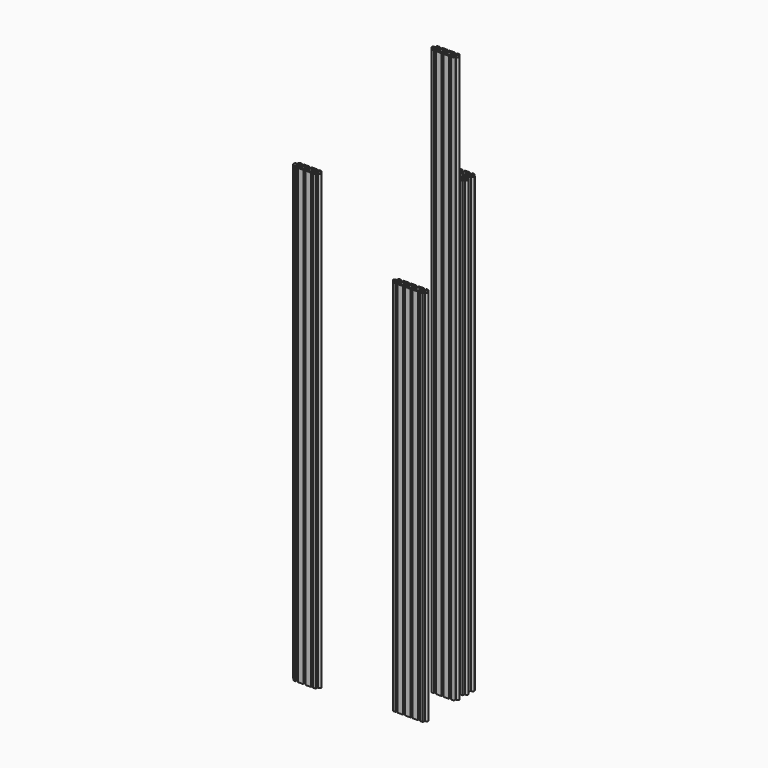
from build123d import *

# Parameters (mm, degrees)
F2_DEPTH = 1500
F3_DEPTH = 1200
F5_DEPTH = 300
F7_DEPTH = 1200
F9_DEPTH = 1000


# Not quite as in the source:
# - ends of sketch curves that miss each other by under 0.0002 mm in the source are joined


with BuildPart() as f2:
    # F0 (on Top) → F2 (new body)
    with BuildSketch(Plane.XY):
        with BuildLine():
            Line((-2.3839193179, -3.6549994873), (0, -3.6549994873))
            Line((0, -3.6549994873), (2.3839193179, -3.6549994873))
            ThreePointArc((2.3839193179, -3.6549994873), (2.5783225274, -3.69366869), (2.7431296106, -3.8037892623))
            Line((2.7431296106, -3.8037892623), (5.8462097795, -6.9068699209))
            ThreePointArc((5.8462097795, -6.9068699209), (5.9563304614, -7.0716774326), (5.9949997993, -7.2660809688))
            Line((5.9949997993, -7.2660809688), (5.9949997993, -7.9920000656))
            ThreePointArc((5.9949997993, -7.9920000656), (5.8462100243, -8.3512103583), (5.4869997316, -8.5000001333))
            Line((5.4869997316, -8.5000001333), (3.1380004184, -8.5000001333))
            ThreePointArc((3.1380004184, -8.5000001333), (2.7787901257, -8.6487899083), (2.6300003507, -9.0080002011))
            Line((2.6300003507, -9.0080002011), (2.6300003507, -9.4920002656))
            ThreePointArc((2.6300003507, -9.4920002656), (2.7787901257, -9.8512105583), (3.1380004184, -10.0000003333))
            Line((3.1380004184, -10.0000003333), (16.8620002483, -10.0000003333))
            ThreePointArc((16.8620002483, -10.0000003333), (17.221210541, -9.8512105583), (17.370000316, -9.4920002656))
            Line((17.370000316, -9.4920002656), (17.370000316, -9.0080002011))
            ThreePointArc((17.370000316, -9.0080002011), (17.221210541, -8.6487899083), (16.8620002483, -8.5000001333))
            Line((16.8620002483, -8.5000001333), (14.5129999351, -8.5000001333))
            ThreePointArc((14.5129999351, -8.5000001333), (14.1537896423, -8.3512103583), (14.0049998673, -7.9920000656))
            Line((14.0049998673, -7.9920000656), (14.0049998673, -7.2660809688))
            ThreePointArc((14.0049998673, -7.2660809688), (14.0436692053, -7.0716774326), (14.1537901423, -6.9068701761))
            Line((14.1537901423, -6.9068701761), (17.2568703009, -3.8037895072))
            ThreePointArc((17.2568703009, -3.8037895072), (17.4216771392, -3.69366869), (17.6160803488, -3.6549994873))
            Line((17.6160803488, -3.6549994873), (22.3839189845, -3.6549994873))
            ThreePointArc((22.3839189845, -3.6549994873), (22.5783221941, -3.69366869), (22.7431292773, -3.8037892623))
            Line((22.7431292773, -3.8037892623), (25.8462104462, -6.9068699209))
            ThreePointArc((25.8462104462, -6.9068699209), (25.9563302634, -7.0716777592), (25.994999466, -7.2660809688))
            Line((25.994999466, -7.2660809688), (25.994999466, -7.9920000656))
            ThreePointArc((25.994999466, -7.9920000656), (25.846209691, -8.3512103583), (25.4869993983, -8.5000001333))
            Line((25.4869993983, -8.5000001333), (23.1380000851, -8.5000001333))
            ThreePointArc((23.1380000851, -8.5000001333), (22.7787897923, -8.6487899083), (22.6300000173, -9.0080002011))
            Line((22.6300000173, -9.0080002011), (22.6300000173, -9.4920002656))
            ThreePointArc((22.6300000173, -9.4920002656), (22.7787897923, -9.8512105583), (23.1380000851, -10.0000003333))
            Line((23.1380000851, -10.0000003333), (28.4999998, -10.0000003333))
            ThreePointArc((28.4999998, -10.0000003333), (29.5606601132, -9.5606604465), (30, -8.5000001333))
            Line((30, -8.5000001333), (30, -3.1618819975))
            ThreePointArc((30, -3.1618819975), (29.7051777422, -2.9096301753), (29.4361827485, -2.6300003507))
            Line((29.4361827485, -2.6300003507), (29.0079998677, -2.6300003507))
            ThreePointArc((29.0079998677, -2.6300003507), (28.648789575, -2.7787901257), (28.4999998, -3.1380004184))
            Line((28.4999998, -3.1380004184), (28.4999998, -5.4869997316))
            ThreePointArc((28.4999998, -5.4869997316), (28.351210025, -5.8462100243), (27.9919997323, -5.9949997993))
            Line((27.9919997323, -5.9949997993), (27.2660806355, -5.9949997993))
            ThreePointArc((27.2660806355, -5.9949997993), (27.0716774259, -5.9563305967), (26.9068703427, -5.8462100243))
            Line((26.9068703427, -5.8462100243), (23.8037891738, -2.7431293658))
            ThreePointArc((23.8037891738, -2.7431293658), (23.6936692213, -2.5783222008), (23.655000154, -2.3839193179))
            Line((23.655000154, -2.3839193179), (23.655000154, 2.3839193179))
            ThreePointArc((23.655000154, 2.3839193179), (23.6936692213, 2.5783222008), (23.803789429, 2.7431291106))
            Line((23.803789429, 2.7431291106), (26.9068705876, 5.8462097795))
            ThreePointArc((26.9068705876, 5.8462097795), (27.0716774259, 5.9563305967), (27.2660806355, 5.9949997993))
            Line((27.2660806355, 5.9949997993), (27.9919997323, 5.9949997993))
            ThreePointArc((27.9919997323, 5.9949997993), (28.351210025, 5.8462100243), (28.4999998, 5.4869997316))
            Line((28.4999998, 5.4869997316), (28.4999998, 3.1380004184))
            ThreePointArc((28.4999998, 3.1380004184), (28.648789575, 2.7787901257), (29.0079998677, 2.6300003507))
            Line((29.0079998677, 2.6300003507), (29.4361827485, 2.6300003507))
            ThreePointArc((29.4361827485, 2.6300003507), (29.7051777422, 2.9096301753), (30, 3.1618819975))
            Line((30, 3.1618819975), (30, 8.5000001333))
            ThreePointArc((30, 8.5000001333), (29.5606601132, 9.5606604465), (28.4999998, 10.0000003333))
            Line((28.4999998, 10.0000003333), (23.1380000851, 10.0000003333))
            ThreePointArc((23.1380000851, 10.0000003333), (22.7787897923, 9.8512105583), (22.6300000173, 9.4920002656))
            Line((22.6300000173, 9.4920002656), (22.6300000173, 9.0080002011))
            ThreePointArc((22.6300000173, 9.0080002011), (22.7787897923, 8.6487899083), (23.1380000851, 8.5000001333))
            Line((23.1380000851, 8.5000001333), (25.4869993983, 8.5000001333))
            ThreePointArc((25.4869993983, 8.5000001333), (25.846209691, 8.3512103583), (25.994999466, 7.9920000656))
            Line((25.994999466, 7.9920000656), (25.994999466, 7.2660809688))
            ThreePointArc((25.994999466, 7.2660809688), (25.9563302634, 7.0716777592), (25.846209691, 6.9068706761))
            Line((25.846209691, 6.9068706761), (22.7431290324, 3.8037895072))
            ThreePointArc((22.7431290324, 3.8037895072), (22.5783221941, 3.69366869), (22.3839189845, 3.6549994873))
            Line((22.3839189845, 3.6549994873), (17.6160803488, 3.6549994873))
            ThreePointArc((17.6160803488, 3.6549994873), (17.4216771392, 3.69366869), (17.2568700561, 3.8037892623))
            Line((17.2568700561, 3.8037892623), (14.1537898872, 6.9068699209))
            ThreePointArc((14.1537898872, 6.9068699209), (14.0436692053, 7.0716774326), (14.0049998673, 7.2660809688))
            Line((14.0049998673, 7.2660809688), (14.0049998673, 7.9920000656))
            ThreePointArc((14.0049998673, 7.9920000656), (14.1537896423, 8.3512103583), (14.5129999351, 8.5000001333))
            Line((14.5129999351, 8.5000001333), (16.8620002483, 8.5000001333))
            ThreePointArc((16.8620002483, 8.5000001333), (17.221210541, 8.6487899083), (17.370000316, 9.0080002011))
            Line((17.370000316, 9.0080002011), (17.370000316, 9.4920002656))
            ThreePointArc((17.370000316, 9.4920002656), (17.221210541, 9.8512105583), (16.8620002483, 10.0000003333))
            Line((16.8620002483, 10.0000003333), (3.1380004184, 10.0000003333))
            ThreePointArc((3.1380004184, 10.0000003333), (2.7787901257, 9.8512105583), (2.6300003507, 9.4920002656))
            Line((2.6300003507, 9.4920002656), (2.6300003507, 9.0080002011))
            ThreePointArc((2.6300003507, 9.0080002011), (2.7787901257, 8.6487899083), (3.1380004184, 8.5000001333))
            Line((3.1380004184, 8.5000001333), (5.4869997316, 8.5000001333))
            ThreePointArc((5.4869997316, 8.5000001333), (5.8462100243, 8.3512103583), (5.9949997993, 7.9920000656))
            Line((5.9949997993, 7.9920000656), (5.9949997993, 7.2660809688))
            ThreePointArc((5.9949997993, 7.2660809688), (5.9563304614, 7.0716774326), (5.8462095243, 6.9068701761))
            Line((5.8462095243, 6.9068701761), (2.7431293658, 3.8037895072))
            ThreePointArc((2.7431293658, 3.8037895072), (2.5783225274, 3.69366869), (2.3839193179, 3.6549994873))
            Line((2.3839193179, 3.6549994873), (0, 3.6549994873))
            Line((0, 3.6549994873), (-2.3839193179, 3.6549994873))
            ThreePointArc((-2.3839193179, 3.6549994873), (-2.5783225274, 3.69366869), (-2.7431296106, 3.8037892623))
            Line((-2.7431296106, 3.8037892623), (-5.8462097795, 6.9068699209))
            ThreePointArc((-5.8462097795, 6.9068699209), (-5.9563304614, 7.0716774326), (-5.9949997993, 7.2660809688))
            Line((-5.9949997993, 7.2660809688), (-5.9949997993, 7.9920000656))
            ThreePointArc((-5.9949997993, 7.9920000656), (-5.8462100243, 8.3512103583), (-5.4869997316, 8.5000001333))
            Line((-5.4869997316, 8.5000001333), (-3.1380004184, 8.5000001333))
            ThreePointArc((-3.1380004184, 8.5000001333), (-2.7787901257, 8.6487899083), (-2.6300003507, 9.0080002011))
            Line((-2.6300003507, 9.0080002011), (-2.6300003507, 9.4920002656))
            ThreePointArc((-2.6300003507, 9.4920002656), (-2.7787901257, 9.8512105583), (-3.1380004184, 10.0000003333))
            Line((-3.1380004184, 10.0000003333), (-16.8620002483, 10.0000003333))
            ThreePointArc((-16.8620002483, 10.0000003333), (-17.221210541, 9.8512105583), (-17.370000316, 9.4920002656))
            Line((-17.370000316, 9.4920002656), (-17.370000316, 9.0080002011))
            ThreePointArc((-17.370000316, 9.0080002011), (-17.221210541, 8.6487899083), (-16.8620002483, 8.5000001333))
            Line((-16.8620002483, 8.5000001333), (-14.5129999351, 8.5000001333))
            ThreePointArc((-14.5129999351, 8.5000001333), (-14.1537896423, 8.3512103583), (-14.0049998673, 7.9920000656))
            Line((-14.0049998673, 7.9920000656), (-14.0049998673, 7.2660809688))
            ThreePointArc((-14.0049998673, 7.2660809688), (-14.0436692053, 7.0716774326), (-14.1537901423, 6.9068701761))
            Line((-14.1537901423, 6.9068701761), (-17.2568703009, 3.8037895072))
            ThreePointArc((-17.2568703009, 3.8037895072), (-17.4216771392, 3.69366869), (-17.6160803488, 3.6549994873))
            Line((-17.6160803488, 3.6549994873), (-22.3839189845, 3.6549994873))
            ThreePointArc((-22.3839189845, 3.6549994873), (-22.5783221941, 3.69366869), (-22.7431292773, 3.8037892623))
            Line((-22.7431292773, 3.8037892623), (-25.8462104462, 6.9068699209))
            ThreePointArc((-25.8462104462, 6.9068699209), (-25.9563302634, 7.0716777592), (-25.994999466, 7.2660809688))
            Line((-25.994999466, 7.2660809688), (-25.994999466, 7.9920000656))
            ThreePointArc((-25.994999466, 7.9920000656), (-25.846209691, 8.3512103583), (-25.4869993983, 8.5000001333))
            Line((-25.4869993983, 8.5000001333), (-23.1380000851, 8.5000001333))
            ThreePointArc((-23.1380000851, 8.5000001333), (-22.7787897923, 8.6487899083), (-22.6300000173, 9.0080002011))
            Line((-22.6300000173, 9.0080002011), (-22.6300000173, 9.4920002656))
            ThreePointArc((-22.6300000173, 9.4920002656), (-22.7787897923, 9.8512105583), (-23.1380000851, 10.0000003333))
            Line((-23.1380000851, 10.0000003333), (-28.4999998, 10.0000003333))
            ThreePointArc((-28.4999998, 10.0000003333), (-29.5606601132, 9.5606604465), (-30, 8.5000001333))
            Line((-30, 8.5000001333), (-30, 3.1618819975))
            ThreePointArc((-30, 3.1618819975), (-29.7051777422, 2.9096301753), (-29.4361827485, 2.6300003507))
            Line((-29.4361827485, 2.6300003507), (-29.0079998677, 2.6300003507))
            ThreePointArc((-29.0079998677, 2.6300003507), (-28.648789575, 2.7787901257), (-28.4999998, 3.1380004184))
            Line((-28.4999998, 3.1380004184), (-28.4999998, 5.4869997316))
            ThreePointArc((-28.4999998, 5.4869997316), (-28.351210025, 5.8462100243), (-27.9919997323, 5.9949997993))
            Line((-27.9919997323, 5.9949997993), (-27.2660806355, 5.9949997993))
            ThreePointArc((-27.2660806355, 5.9949997993), (-27.0716774259, 5.9563305967), (-26.9068703427, 5.8462100243))
            Line((-26.9068703427, 5.8462100243), (-23.8037891738, 2.7431293658))
            ThreePointArc((-23.8037891738, 2.7431293658), (-23.6936692213, 2.5783222008), (-23.655000154, 2.3839193179))
            Line((-23.655000154, 2.3839193179), (-23.655000154, -2.3839193179))
            ThreePointArc((-23.655000154, -2.3839193179), (-23.6936692213, -2.5783222008), (-23.803789429, -2.7431291106))
            Line((-23.803789429, -2.7431291106), (-26.9068705876, -5.8462097795))
            ThreePointArc((-26.9068705876, -5.8462097795), (-27.0716774259, -5.9563305967), (-27.2660806355, -5.9949997993))
            Line((-27.2660806355, -5.9949997993), (-27.9919997323, -5.9949997993))
            ThreePointArc((-27.9919997323, -5.9949997993), (-28.351210025, -5.8462100243), (-28.4999998, -5.4869997316))
            Line((-28.4999998, -5.4869997316), (-28.4999998, -3.1380004184))
            ThreePointArc((-28.4999998, -3.1380004184), (-28.648789575, -2.7787901257), (-29.0079998677, -2.6300003507))
            Line((-29.0079998677, -2.6300003507), (-29.4361827485, -2.6300003507))
            ThreePointArc((-29.4361827485, -2.6300003507), (-29.7051777422, -2.9096301753), (-30, -3.1618819975))
            Line((-30, -3.1618819975), (-30, -8.5000001333))
            ThreePointArc((-30, -8.5000001333), (-29.5606601132, -9.5606604465), (-28.4999998, -10.0000003333))
            Line((-28.4999998, -10.0000003333), (-23.1380000851, -10.0000003333))
            ThreePointArc((-23.1380000851, -10.0000003333), (-22.7787897923, -9.8512105583), (-22.6300000173, -9.4920002656))
            Line((-22.6300000173, -9.4920002656), (-22.6300000173, -9.0080002011))
            ThreePointArc((-22.6300000173, -9.0080002011), (-22.7787897923, -8.6487899083), (-23.1380000851, -8.5000001333))
            Line((-23.1380000851, -8.5000001333), (-25.4869993983, -8.5000001333))
            ThreePointArc((-25.4869993983, -8.5000001333), (-25.846209691, -8.3512103583), (-25.994999466, -7.9920000656))
            Line((-25.994999466, -7.9920000656), (-25.994999466, -7.2660809688))
            ThreePointArc((-25.994999466, -7.2660809688), (-25.9563302634, -7.0716777592), (-25.846209691, -6.9068706761))
            Line((-25.846209691, -6.9068706761), (-22.7431290324, -3.8037895072))
            ThreePointArc((-22.7431290324, -3.8037895072), (-22.5783221941, -3.69366869), (-22.3839189845, -3.6549994873))
            Line((-22.3839189845, -3.6549994873), (-17.6160803488, -3.6549994873))
            ThreePointArc((-17.6160803488, -3.6549994873), (-17.4216771392, -3.69366869), (-17.2568700561, -3.8037892623))
            Line((-17.2568700561, -3.8037892623), (-14.1537898872, -6.9068699209))
            ThreePointArc((-14.1537898872, -6.9068699209), (-14.0436692053, -7.0716774326), (-14.0049998673, -7.2660809688))
            Line((-14.0049998673, -7.2660809688), (-14.0049998673, -7.9920000656))
            ThreePointArc((-14.0049998673, -7.9920000656), (-14.1537896423, -8.3512103583), (-14.5129999351, -8.5000001333))
            Line((-14.5129999351, -8.5000001333), (-16.8620002483, -8.5000001333))
            ThreePointArc((-16.8620002483, -8.5000001333), (-17.221210541, -8.6487899083), (-17.370000316, -9.0080002011))
            Line((-17.370000316, -9.0080002011), (-17.370000316, -9.4920002656))
            ThreePointArc((-17.370000316, -9.4920002656), (-17.221210541, -9.8512105583), (-16.8620002483, -10.0000003333))
            Line((-16.8620002483, -10.0000003333), (-3.1380004184, -10.0000003333))
            ThreePointArc((-3.1380004184, -10.0000003333), (-2.7787901257, -9.8512105583), (-2.6300003507, -9.4920002656))
            Line((-2.6300003507, -9.4920002656), (-2.6300003507, -9.0080002011))
            ThreePointArc((-2.6300003507, -9.0080002011), (-2.7787901257, -8.6487899083), (-3.1380004184, -8.5000001333))
            Line((-3.1380004184, -8.5000001333), (-5.4869997316, -8.5000001333))
            ThreePointArc((-5.4869997316, -8.5000001333), (-5.8462100243, -8.3512103583), (-5.9949997993, -7.9920000656))
            Line((-5.9949997993, -7.9920000656), (-5.9949997993, -7.2660809688))
            ThreePointArc((-5.9949997993, -7.2660809688), (-5.9563304614, -7.0716774326), (-5.8462095243, -6.9068701761))
            Line((-5.8462095243, -6.9068701761), (-2.7431293658, -3.8037895072))
            ThreePointArc((-2.7431293658, -3.8037895072), (-2.5783225274, -3.69366869), (-2.3839193179, -3.6549994873))
        make_face()
        with BuildLine():
            ThreePointArc((-19.1960237766, 1.9351333112), (-18.6435327415, 2.5059383489), (-17.8750993466, 2.3045063441))
            Line((-17.8750993466, 2.3045063441), (-17.6954943594, 2.1249012833))
            ThreePointArc((-17.6954943594, 2.1249012833), (-17.494062187, 1.3564683929), (-18.064866412, 0.803977121))
            ThreePointArc((-18.064866412, 0.803977121), (-17.9044993873, 0), (-18.0648660769, -0.803977245))
            ThreePointArc((-18.0648660769, -0.803977245), (-17.494062187, -1.3564683929), (-17.6954943226, -2.1249013201))
            Line((-17.6954943226, -2.1249013201), (-17.8750993833, -2.3045063073))
            ThreePointArc((-17.8750993833, -2.3045063073), (-18.6435327415, -2.5059383489), (-19.1960237766, -1.9351333112))
            ThreePointArc((-19.1960237766, -1.9351333112), (-20.0000001284, -2.0955002794), (-20.8039769117, -1.9351335898))
            ThreePointArc((-20.8039769117, -1.9351335898), (-21.3564675919, -2.5059383489), (-22.1249009868, -2.3045063441))
            Line((-22.1249009868, -2.3045063441), (-22.3045059739, -2.1249012833))
            ThreePointArc((-22.3045059739, -2.1249012833), (-22.5059380156, -1.3564679252), (-21.9351329778, -0.8039768901))
            ThreePointArc((-21.9351329778, -0.8039768901), (-22.0954999461, 0), (-21.9351332565, 0.803977245))
            ThreePointArc((-21.9351332565, 0.803977245), (-22.5059380156, 1.3564679252), (-22.3045060107, 2.1249013201))
            Line((-22.3045060107, 2.1249013201), (-22.12490095, 2.3045063073))
            ThreePointArc((-22.12490095, 2.3045063073), (-21.3564675919, 2.5059383489), (-20.8039765567, 1.9351333112))
            ThreePointArc((-20.8039765567, 1.9351333112), (-20.0000001284, 2.0955002794), (-19.1960237766, 1.9351333112))
        make_face(mode=Mode.SUBTRACT)
        with BuildLine():
            ThreePointArc((-3.8037892623, 2.7431296106), (-3.69366869, 2.5783225274), (-3.6549994873, 2.3839193179))
            Line((-3.6549994873, 2.3839193179), (-3.6549994873, -2.3839193179))
            ThreePointArc((-3.6549994873, -2.3839193179), (-3.69366869, -2.5783225274), (-3.8037892623, -2.7431296106))
            Line((-3.8037892623, -2.7431296106), (-7.3462099795, -6.2855498381))
            ThreePointArc((-7.3462099795, -6.2855498381), (-7.4563307967, -6.4503566764), (-7.4949999993, -6.644759886))
            Line((-7.4949999993, -6.644759886), (-7.4949999993, -7.9920000656))
            ThreePointArc((-7.4949999993, -7.9920000656), (-7.6437897743, -8.3512103583), (-8.0030000671, -8.5000001333))
            Line((-8.0030000671, -8.5000001333), (-11.9969995996, -8.5000001333))
            ThreePointArc((-11.9969995996, -8.5000001333), (-12.3562098923, -8.3512103583), (-12.5049996673, -7.9920000656))
            Line((-12.5049996673, -7.9920000656), (-12.5049996673, -6.644759886))
            ThreePointArc((-12.5049996673, -6.644759886), (-12.54366887, -6.4503566764), (-12.6537894423, -6.2855495932))
            Line((-12.6537894423, -6.2855495932), (-16.1962101595, -2.7431293658))
            ThreePointArc((-16.1962101595, -2.7431293658), (-16.3063309767, -2.5783225274), (-16.3450001793, -2.3839193179))
            Line((-16.3450001793, -2.3839193179), (-16.3450001793, 2.3839193179))
            ThreePointArc((-16.3450001793, 2.3839193179), (-16.3063309767, 2.5783225274), (-16.1962104043, 2.7431296106))
            Line((-16.1962104043, 2.7431296106), (-12.6537896872, 6.2855498381))
            ThreePointArc((-12.6537896872, 6.2855498381), (-12.54366887, 6.4503566764), (-12.5049996673, 6.644759886))
            Line((-12.5049996673, 6.644759886), (-12.5049996673, 7.9920000656))
            ThreePointArc((-12.5049996673, 7.9920000656), (-12.3562098923, 8.3512103583), (-11.9969995996, 8.5000001333))
            Line((-11.9969995996, 8.5000001333), (-8.0030000671, 8.5000001333))
            ThreePointArc((-8.0030000671, 8.5000001333), (-7.6437897743, 8.3512103583), (-7.4949999993, 7.9920000656))
            Line((-7.4949999993, 7.9920000656), (-7.4949999993, 6.644759886))
            ThreePointArc((-7.4949999993, 6.644759886), (-7.4563307967, 6.4503566764), (-7.3462102243, 6.2855495932))
            Line((-7.3462102243, 6.2855495932), (-3.8037892623, 2.7431296106))
        make_face(mode=Mode.SUBTRACT)
        with BuildLine():
            ThreePointArc((-2.1249013201, 2.3045063441), (-1.3564679252, 2.5059383489), (-0.8039768901, 1.9351333112))
            ThreePointArc((-0.8039768901, 1.9351333112), (-0.4099075767, 2.0550175667), (0, 2.0955002794))
            ThreePointArc((0, 2.0955002794), (0.4099075767, 2.0550175667), (0.803977245, 1.9351335898))
            ThreePointArc((0.803977245, 1.9351335898), (1.3564679252, 2.5059383489), (2.1249013201, 2.3045063441))
            Line((2.1249013201, 2.3045063441), (2.3045063073, 2.1249012833))
            ThreePointArc((2.3045063073, 2.1249012833), (2.5059383489, 1.3564679252), (1.9351333112, 0.8039768901))
            ThreePointArc((1.9351333112, 0.8039768901), (2.0955002794, 0), (1.9351335898, -0.803977245))
            ThreePointArc((1.9351335898, -0.803977245), (2.5059383489, -1.3564679252), (2.3045063441, -2.1249013201))
            Line((2.3045063441, -2.1249013201), (2.1249012833, -2.3045063073))
            ThreePointArc((2.1249012833, -2.3045063073), (1.3564679252, -2.5059383489), (0.8039768901, -1.9351333112))
            ThreePointArc((0.8039768901, -1.9351333112), (0.4099075767, -2.0550175667), (0, -2.0955002794))
            ThreePointArc((0, -2.0955002794), (-0.4099075767, -2.0550175667), (-0.803977245, -1.9351335898))
            ThreePointArc((-0.803977245, -1.9351335898), (-1.3564679252, -2.5059383489), (-2.1249013201, -2.3045063441))
            Line((-2.1249013201, -2.3045063441), (-2.3045063073, -2.1249012833))
            ThreePointArc((-2.3045063073, -2.1249012833), (-2.5059383489, -1.3564679252), (-1.9351333112, -0.8039768901))
            ThreePointArc((-1.9351333112, -0.8039768901), (-2.0955002794, 0), (-1.9351335898, 0.803977245))
            ThreePointArc((-1.9351335898, 0.803977245), (-2.5059383489, 1.3564679252), (-2.3045063441, 2.1249013201))
            Line((-2.3045063441, 2.1249013201), (-2.1249013201, 2.3045063441))
        make_face(mode=Mode.SUBTRACT)
        with BuildLine():
            Line((3.6549994873, -2.3839193179), (3.6549994873, 2.3839193179))
            ThreePointArc((3.6549994873, 2.3839193179), (3.69366869, 2.5783225274), (3.8037892623, 2.7431296106))
            Line((3.8037892623, 2.7431296106), (7.3462099795, 6.2855498381))
            ThreePointArc((7.3462099795, 6.2855498381), (7.4563307967, 6.4503566764), (7.4949999993, 6.644759886))
            Line((7.4949999993, 6.644759886), (7.4949999993, 7.9920000656))
            ThreePointArc((7.4949999993, 7.9920000656), (7.6437897743, 8.3512103583), (8.0030000671, 8.5000001333))
            Line((8.0030000671, 8.5000001333), (11.9969995996, 8.5000001333))
            ThreePointArc((11.9969995996, 8.5000001333), (12.3562098923, 8.3512103583), (12.5049996673, 7.9920000656))
            Line((12.5049996673, 7.9920000656), (12.5049996673, 6.644759886))
            ThreePointArc((12.5049996673, 6.644759886), (12.54366887, 6.4503566764), (12.6537894423, 6.2855495932))
            Line((12.6537894423, 6.2855495932), (16.1962101595, 2.7431293658))
            ThreePointArc((16.1962101595, 2.7431293658), (16.3063309767, 2.5783225274), (16.3450001793, 2.3839193179))
            Line((16.3450001793, 2.3839193179), (16.3450001793, -2.3839193179))
            ThreePointArc((16.3450001793, -2.3839193179), (16.3063309767, -2.5783225274), (16.1962104043, -2.7431296106))
            Line((16.1962104043, -2.7431296106), (12.6537896872, -6.2855498381))
            ThreePointArc((12.6537896872, -6.2855498381), (12.54366887, -6.4503566764), (12.5049996673, -6.644759886))
            Line((12.5049996673, -6.644759886), (12.5049996673, -7.9920000656))
            ThreePointArc((12.5049996673, -7.9920000656), (12.3562098923, -8.3512103583), (11.9969995996, -8.5000001333))
            Line((11.9969995996, -8.5000001333), (8.0030000671, -8.5000001333))
            ThreePointArc((8.0030000671, -8.5000001333), (7.6437897743, -8.3512103583), (7.4949999993, -7.9920000656))
            Line((7.4949999993, -7.9920000656), (7.4949999993, -6.644759886))
            ThreePointArc((7.4949999993, -6.644759886), (7.4563307967, -6.4503566764), (7.3462102243, -6.2855495932))
            Line((7.3462102243, -6.2855495932), (3.8037895072, -2.7431293658))
            ThreePointArc((3.8037895072, -2.7431293658), (3.69366869, -2.5783225274), (3.6549994873, -2.3839193179))
        make_face(mode=Mode.SUBTRACT)
        with BuildLine():
            Line((17.6954943594, 2.1249012833), (17.8750993833, 2.3045063073))
            ThreePointArc((17.8750993833, 2.3045063073), (18.6435327415, 2.5059383489), (19.1960237766, 1.9351333112))
            ThreePointArc((19.1960237766, 1.9351333112), (20.0000001284, 2.0955002794), (20.8039769117, 1.9351335898))
            ThreePointArc((20.8039769117, 1.9351335898), (21.3564675919, 2.5059383489), (22.1249009868, 2.3045063441))
            Line((22.1249009868, 2.3045063441), (22.3045059739, 2.1249012833))
            ThreePointArc((22.3045059739, 2.1249012833), (22.5059380156, 1.3564679252), (21.9351329778, 0.8039768901))
            ThreePointArc((21.9351329778, 0.8039768901), (22.0954999461, 0), (21.9351332565, -0.803977245))
            ThreePointArc((21.9351332565, -0.803977245), (22.5059380156, -1.3564679252), (22.3045060107, -2.1249013201))
            Line((22.3045060107, -2.1249013201), (22.12490095, -2.3045063073))
            ThreePointArc((22.12490095, -2.3045063073), (21.3564675919, -2.5059383489), (20.8039765567, -1.9351333112))
            ThreePointArc((20.8039765567, -1.9351333112), (20.0000001284, -2.0955002794), (19.1960232744, -1.9351339441))
            ThreePointArc((19.1960232744, -1.9351339441), (18.6435327415, -2.5059383489), (17.8750993466, -2.3045063441))
            Line((17.8750993466, -2.3045063441), (17.6954943594, -2.1249012833))
            ThreePointArc((17.6954943594, -2.1249012833), (17.494062187, -1.3564683929), (18.064866412, -0.803977121))
            ThreePointArc((18.064866412, -0.803977121), (17.9044993873, 0), (18.0648660769, 0.803977245))
            ThreePointArc((18.0648660769, 0.803977245), (17.494062187, 1.3564683929), (17.6954943594, 2.1249012833))
        make_face(mode=Mode.SUBTRACT)
        with BuildLine():
            ThreePointArc((-30, 3.1618819975), (-36.45000186, 0), (-30, -3.1618819975))
            Line((-30, -3.1618819975), (-30, -3.1380004184))
            ThreePointArc((-30, -3.1380004184), (-29.851210225, -2.7787901257), (-29.4919999323, -2.6300003507))
            Line((-29.4919999323, -2.6300003507), (-29.4361827485, -2.6300003507))
            ThreePointArc((-29.4361827485, -2.6300003507), (-28.7046521983, -1.4044088341), (-28.4500007933, 0))
            ThreePointArc((-28.4500007933, 0), (-28.7046521983, 1.4044088341), (-29.4361827485, 2.6300003507))
            Line((-29.4361827485, 2.6300003507), (-29.4919999323, 2.6300003507))
            ThreePointArc((-29.4919999323, 2.6300003507), (-29.851210225, 2.7787901257), (-30, 3.1380004184))
            Line((-30, 3.1380004184), (-30, 3.1618819975))
        make_face()
        with BuildLine():
            Line((-30, -3.1380004184), (-30, -3.1618819975))
            ThreePointArc((-30, -3.1618819975), (-29.7051777422, -2.9096301753), (-29.4361827485, -2.6300003507))
            Line((-29.4361827485, -2.6300003507), (-29.4919999323, -2.6300003507))
            ThreePointArc((-29.4919999323, -2.6300003507), (-29.851210225, -2.7787901257), (-30, -3.1380004184))
        make_face()
        with BuildLine():
            ThreePointArc((29.4361827485, -2.6300003507), (29.7051777422, -2.9096301753), (30, -3.1618819975))
            Line((30, -3.1618819975), (30, -3.1380004184))
            ThreePointArc((30, -3.1380004184), (29.851210225, -2.7787901257), (29.4919999323, -2.6300003507))
            Line((29.4919999323, -2.6300003507), (29.4361827485, -2.6300003507))
        make_face()
        with BuildLine():
            Line((30, -3.1380004184), (30, -3.1618819975))
            ThreePointArc((30, -3.1618819975), (34.2106826796, -3.5916577565), (36.45000186, 0))
            ThreePointArc((36.45000186, 0), (34.2106826796, 3.5916577565), (30, 3.1618819975))
            Line((30, 3.1618819975), (30, 3.1380004184))
            ThreePointArc((30, 3.1380004184), (29.851210225, 2.7787901257), (29.4919999323, 2.6300003507))
            Line((29.4919999323, 2.6300003507), (29.4361827485, 2.6300003507))
            ThreePointArc((29.4361827485, 2.6300003507), (28.4500007933, 0), (29.4361827485, -2.6300003507))
            Line((29.4361827485, -2.6300003507), (29.4919999323, -2.6300003507))
            ThreePointArc((29.4919999323, -2.6300003507), (29.851210225, -2.7787901257), (30, -3.1380004184))
        make_face()
        with BuildLine():
            ThreePointArc((-29.4361827485, 2.6300003507), (-29.7051777422, 2.9096301753), (-30, 3.1618819975))
            Line((-30, 3.1618819975), (-30, 3.1380004184))
            ThreePointArc((-30, 3.1380004184), (-29.851210225, 2.7787901257), (-29.4919999323, 2.6300003507))
            Line((-29.4919999323, 2.6300003507), (-29.4361827485, 2.6300003507))
        make_face()
        with BuildLine():
            ThreePointArc((30, 3.1618819975), (29.7051777422, 2.9096301753), (29.4361827485, 2.6300003507))
            Line((29.4361827485, 2.6300003507), (29.4919999323, 2.6300003507))
            ThreePointArc((29.4919999323, 2.6300003507), (29.851210225, 2.7787901257), (30, 3.1380004184))
            Line((30, 3.1380004184), (30, 3.1618819975))
        make_face()
    extrude(amount=F2_DEPTH)


with BuildPart() as f3:
    # F1 (on Top) → F3 (new body)
    with BuildSketch(Plane.XY):
        with BuildLine():
            Line((-29.99999975, 46.8381304789), (-29.99999975, 38.5000130125))
            Line((-29.99999975, 38.5000130125), (-29.99999975, 33.1618949211))
            ThreePointArc((-29.99999975, 33.1618949211), (-29.705177012, 32.9096426457), (-29.4361816305, 32.6300122787))
            Line((-29.4361816305, 32.6300122787), (-29.007999626, 32.6300122787))
            ThreePointArc((-29.007999626, 32.6300122787), (-28.6487893363, 32.7788020525), (-28.4999995625, 33.1380123423))
            Line((-28.4999995625, 33.1380123423), (-28.4999995625, 35.4870126359))
            ThreePointArc((-28.4999995625, 35.4870126359), (-28.3512097887, 35.8462229256), (-27.991999499, 35.9950126994))
            Line((-27.991999499, 35.9950126994), (-27.2660804083, 35.9950126994))
            ThreePointArc((-27.2660804083, 35.9950126994), (-27.0716772003, 35.9563434971), (-26.9068701185, 35.8462229256))
            Line((-26.9068701185, 35.8462229256), (-23.8037889755, 32.7431422929))
            ThreePointArc((-23.8037889755, 32.7431422929), (-23.6936690239, 32.5783351293), (-23.6549999569, 32.383932248))
            Line((-23.6549999569, 32.383932248), (-23.6549999569, 27.616093652))
            ThreePointArc((-23.6549999569, 27.616093652), (-23.6936690239, 27.4216907707), (-23.8037892306, 27.2568838623))
            Line((-23.8037892306, 27.2568838623), (-26.9068703634, 24.1538022192))
            ThreePointArc((-26.9068703634, 24.1538022192), (-27.071677527, 24.0436822676), (-27.2660804083, 24.0050132006))
            Line((-27.2660804083, 24.0050132006), (-27.991999499, 24.0050132006))
            ThreePointArc((-27.991999499, 24.0050132006), (-28.3512097887, 24.1538029744), (-28.4999995625, 24.5130132641))
            Line((-28.4999995625, 24.5130132641), (-28.4999995625, 26.8620125578))
            ThreePointArc((-28.4999995625, 26.8620125578), (-28.6487893363, 27.2212228475), (-29.007999626, 27.3700126213))
            Line((-29.007999626, 27.3700126213), (-29.4361825032, 27.3700126213))
            ThreePointArc((-29.4361825032, 27.3700126213), (-29.7051774947, 27.090382799), (-29.99999975, 26.8381309789))
            Line((-29.99999975, 26.8381309789), (-29.99999975, 21.5000128875))
            ThreePointArc((-29.99999975, 21.5000128875), (-29.5606598669, 20.4393525831), (-28.4999995625, 20.0000127))
            Line((-28.4999995625, 20.0000127), (-23.1379998922, 20.0000127))
            ThreePointArc((-23.1379998922, 20.0000127), (-22.7787896025, 20.1488024738), (-22.6299998287, 20.5080127635))
            Line((-22.6299998287, 20.5080127635), (-22.6299998287, 20.992012824))
            ThreePointArc((-22.6299998287, 20.992012824), (-22.7787896025, 21.3512231137), (-23.1379998922, 21.5000128875))
            Line((-23.1379998922, 21.5000128875), (-25.4869991859, 21.5000128875))
            ThreePointArc((-25.4869991859, 21.5000128875), (-25.8462094756, 21.6488026613), (-25.9949992494, 22.008012951))
            Line((-25.9949992494, 22.008012951), (-25.9949992494, 22.7339320417))
            ThreePointArc((-25.9949992494, 22.7339320417), (-25.9563301824, 22.928334923), (-25.8462099756, 23.0931418315))
            Line((-25.8462099756, 23.0931418315), (-22.7431288429, 26.1962234745))
            ThreePointArc((-22.7431288429, 26.1962234745), (-22.5783216793, 26.3063434261), (-22.383918798, 26.3450124931))
            Line((-22.383918798, 26.3450124931), (-17.616080202, 26.3450124931))
            ThreePointArc((-17.616080202, 26.3450124931), (-17.4216773207, 26.3063434261), (-17.2568704123, 26.1962232194))
            Line((-17.2568704123, 26.1962232194), (-14.1537897692, 23.0931420866))
            ThreePointArc((-14.1537897692, 23.0931420866), (-14.0436689529, 22.9283352497), (-14.0049997506, 22.7339320417))
            Line((-14.0049997506, 22.7339320417), (-14.0049997506, 22.008012951))
            ThreePointArc((-14.0049997506, 22.008012951), (-14.1537895244, 21.6488026613), (-14.5129998141, 21.5000128875))
            Line((-14.5129998141, 21.5000128875), (-16.8620001078, 21.5000128875))
            ThreePointArc((-16.8620001078, 21.5000128875), (-17.2212103975, 21.3512231137), (-17.3700001713, 20.992012824))
            Line((-17.3700001713, 20.992012824), (-17.3700001713, 20.5080127635))
            ThreePointArc((-17.3700001713, 20.5080127635), (-17.2212103975, 20.1488024738), (-16.8620001078, 20.0000127))
            Line((-16.8620001078, 20.0000127), (-3.1380003923, 20.0000127))
            ThreePointArc((-3.1380003923, 20.0000127), (-2.7787901025, 20.1488024738), (-2.6300003288, 20.5080127635))
            Line((-2.6300003288, 20.5080127635), (-2.6300003288, 20.992012824))
            ThreePointArc((-2.6300003288, 20.992012824), (-2.7787901025, 21.3512231137), (-3.1380003923, 21.5000128875))
            Line((-3.1380003923, 21.5000128875), (-5.4869996859, 21.5000128875))
            ThreePointArc((-5.4869996859, 21.5000128875), (-5.8462099756, 21.6488026613), (-5.9949997494, 22.008012951))
            Line((-5.9949997494, 22.008012951), (-5.9949997494, 22.7339320417))
            ThreePointArc((-5.9949997494, 22.7339320417), (-5.9563305471, 22.9283352497), (-5.8462099756, 23.0931423315))
            Line((-5.8462099756, 23.0931423315), (-2.7431293429, 26.1962234745))
            ThreePointArc((-2.7431293429, 26.1962234745), (-2.5783221793, 26.3063434261), (-2.383919298, 26.3450124931))
            Line((-2.383919298, 26.3450124931), (0, 26.3450124931))
            Line((0, 26.3450124931), (2.383919298, 26.3450124931))
            ThreePointArc((2.383919298, 26.3450124931), (2.5783221793, 26.3063434261), (2.7431290877, 26.1962232194))
            Line((2.7431290877, 26.1962232194), (5.8462097308, 23.0931420866))
            ThreePointArc((5.8462097308, 23.0931420866), (5.9563305471, 22.9283352497), (5.9949997494, 22.7339320417))
            Line((5.9949997494, 22.7339320417), (5.9949997494, 22.008012951))
            ThreePointArc((5.9949997494, 22.008012951), (5.8462099756, 21.6488026613), (5.4869996859, 21.5000128875))
            Line((5.4869996859, 21.5000128875), (3.1380003923, 21.5000128875))
            ThreePointArc((3.1380003923, 21.5000128875), (2.7787901025, 21.3512231137), (2.6300003288, 20.992012824))
            Line((2.6300003288, 20.992012824), (2.6300003288, 20.5080127635))
            ThreePointArc((2.6300003288, 20.5080127635), (2.7787901025, 20.1488024738), (3.1380003923, 20.0000127))
            Line((3.1380003923, 20.0000127), (16.8620001078, 20.0000127))
            ThreePointArc((16.8620001078, 20.0000127), (17.2212103975, 20.1488024738), (17.3700001713, 20.5080127635))
            Line((17.3700001713, 20.5080127635), (17.3700001713, 20.992012824))
            ThreePointArc((17.3700001713, 20.992012824), (17.2212103975, 21.3512231137), (16.8620001078, 21.5000128875))
            Line((16.8620001078, 21.5000128875), (14.5129998141, 21.5000128875))
            ThreePointArc((14.5129998141, 21.5000128875), (14.1537895244, 21.6488026613), (14.0049997506, 22.008012951))
            Line((14.0049997506, 22.008012951), (14.0049997506, 22.7339320417))
            ThreePointArc((14.0049997506, 22.7339320417), (14.0436689529, 22.9283352497), (14.1537895244, 23.0931423315))
            Line((14.1537895244, 23.0931423315), (17.2568701571, 26.1962234745))
            ThreePointArc((17.2568701571, 26.1962234745), (17.4216773207, 26.3063434261), (17.616080202, 26.3450124931))
            Line((17.616080202, 26.3450124931), (22.383918798, 26.3450124931))
            ThreePointArc((22.383918798, 26.3450124931), (22.5783216793, 26.3063434261), (22.7431285877, 26.1962232194))
            Line((22.7431285877, 26.1962232194), (25.8462102308, 23.0931420866))
            ThreePointArc((25.8462102308, 23.0931420866), (25.9563301824, 22.928334923), (25.9949992494, 22.7339320417))
            Line((25.9949992494, 22.7339320417), (25.9949992494, 22.008012951))
            ThreePointArc((25.9949992494, 22.008012951), (25.8462094756, 21.6488026613), (25.4869991859, 21.5000128875))
            Line((25.4869991859, 21.5000128875), (23.1379998922, 21.5000128875))
            ThreePointArc((23.1379998922, 21.5000128875), (22.7787896025, 21.3512231137), (22.6299998287, 20.992012824))
            Line((22.6299998287, 20.992012824), (22.6299998287, 20.5080127635))
            ThreePointArc((22.6299998287, 20.5080127635), (22.7787896025, 20.1488024738), (23.1379998922, 20.0000127))
            Line((23.1379998922, 20.0000127), (28.4999995625, 20.0000127))
            ThreePointArc((28.4999995625, 20.0000127), (29.5606598669, 20.4393525831), (29.99999975, 21.5000128875))
            Line((29.99999975, 21.5000128875), (29.99999975, 26.8381309789))
            ThreePointArc((29.99999975, 26.8381309789), (29.7051774947, 27.090382799), (29.4361825032, 27.3700126213))
            Line((29.4361825032, 27.3700126213), (29.007999626, 27.3700126213))
            ThreePointArc((29.007999626, 27.3700126213), (28.6487893363, 27.2212228475), (28.4999995625, 26.8620125578))
            Line((28.4999995625, 26.8620125578), (28.4999995625, 24.5130132641))
            ThreePointArc((28.4999995625, 24.5130132641), (28.3512097887, 24.1538029744), (27.991999499, 24.0050132006))
            Line((27.991999499, 24.0050132006), (27.2660804083, 24.0050132006))
            ThreePointArc((27.2660804083, 24.0050132006), (27.071677527, 24.0436822676), (26.9068706185, 24.1538024744))
            Line((26.9068706185, 24.1538024744), (23.8037889755, 27.2568836071))
            ThreePointArc((23.8037889755, 27.2568836071), (23.6936690239, 27.4216907707), (23.6549999569, 27.616093652))
            Line((23.6549999569, 27.616093652), (23.6549999569, 32.383932248))
            ThreePointArc((23.6549999569, 32.383932248), (23.6936690239, 32.5783351293), (23.8037892306, 32.7431420377))
            Line((23.8037892306, 32.7431420377), (26.9068703634, 35.8462226808))
            ThreePointArc((26.9068703634, 35.8462226808), (27.0716772003, 35.9563434971), (27.2660804083, 35.9950126994))
            Line((27.2660804083, 35.9950126994), (27.991999499, 35.9950126994))
            ThreePointArc((27.991999499, 35.9950126994), (28.3512097887, 35.8462229256), (28.4999995625, 35.4870126359))
            Line((28.4999995625, 35.4870126359), (28.4999995625, 33.1380123423))
            ThreePointArc((28.4999995625, 33.1380123423), (28.6487893363, 32.7788020525), (29.007999626, 32.6300122788))
            Line((29.007999626, 32.6300122788), (29.4361816305, 32.6300122787))
            ThreePointArc((29.4361816305, 32.6300122787), (29.705177012, 32.9096426457), (29.99999975, 33.1618949211))
            Line((29.99999975, 33.1618949211), (29.99999975, 38.5000130125))
            Line((29.99999975, 38.5000130125), (29.99999975, 46.8381304789))
            ThreePointArc((29.99999975, 46.8381304789), (29.7051774947, 47.090382299), (29.4361825032, 47.3700121212))
            Line((29.4361825032, 47.3700121212), (29.007999626, 47.3700121212))
            ThreePointArc((29.007999626, 47.3700121212), (28.6487893363, 47.2212223475), (28.4999995625, 46.8620120577))
            Line((28.4999995625, 46.8620120577), (28.4999995625, 44.5130127641))
            ThreePointArc((28.4999995625, 44.5130127641), (28.3512097887, 44.1538024744), (27.991999499, 44.0050127006))
            Line((27.991999499, 44.0050127006), (27.2660804083, 44.0050127006))
            ThreePointArc((27.2660804083, 44.0050127006), (27.0716772003, 44.0436819029), (26.9068701185, 44.1538024744))
            Line((26.9068701185, 44.1538024744), (23.8037889755, 47.2568831071))
            ThreePointArc((23.8037889755, 47.2568831071), (23.6936690239, 47.4216902707), (23.6549999569, 47.616093152))
            Line((23.6549999569, 47.616093152), (23.6549999569, 52.383931748))
            ThreePointArc((23.6549999569, 52.383931748), (23.6936690239, 52.5783346293), (23.8037892306, 52.7431415377))
            Line((23.8037892306, 52.7431415377), (26.9068703634, 55.8462221808))
            ThreePointArc((26.9068703634, 55.8462221808), (27.0716772003, 55.9563429971), (27.2660804083, 55.9950121994))
            Line((27.2660804083, 55.9950121994), (27.991999499, 55.9950121994))
            ThreePointArc((27.991999499, 55.9950121994), (28.3512097887, 55.8462224256), (28.4999995625, 55.4870121359))
            Line((28.4999995625, 55.4870121359), (28.4999995625, 53.1380128423))
            ThreePointArc((28.4999995625, 53.1380128423), (28.6487893363, 52.7788025525), (29.007999626, 52.6300127788))
            Line((29.007999626, 52.6300127788), (29.4361825032, 52.6300127788))
            ThreePointArc((29.4361825032, 52.6300127788), (29.7051774947, 52.909642601), (29.99999975, 53.1618944211))
            Line((29.99999975, 53.1618944211), (29.99999975, 58.5000125125))
            ThreePointArc((29.99999975, 58.5000125125), (29.5606598669, 59.5606728169), (28.4999995625, 60.0000127))
            Line((28.4999995625, 60.0000127), (23.1379998922, 60.0000127))
            ThreePointArc((23.1379998922, 60.0000127), (22.7787896025, 59.8512229262), (22.6299998287, 59.4920126365))
            Line((22.6299998287, 59.4920126365), (22.6299998287, 59.008012576))
            ThreePointArc((22.6299998287, 59.008012576), (22.7787896025, 58.6488022863), (23.1379998922, 58.5000125125))
            Line((23.1379998922, 58.5000125125), (25.4869991859, 58.5000125125))
            ThreePointArc((25.4869991859, 58.5000125125), (25.8462094756, 58.3512227387), (25.9949992494, 57.992012449))
            Line((25.9949992494, 57.992012449), (25.9949992494, 57.2660933583))
            ThreePointArc((25.9949992494, 57.2660933583), (25.9563300471, 57.0716901503), (25.8462094756, 56.9068830685))
            Line((25.8462094756, 56.9068830685), (22.7431288429, 53.8038019255))
            ThreePointArc((22.7431288429, 53.8038019255), (22.5783220059, 53.6936811092), (22.383918798, 53.6550119069))
            Line((22.383918798, 53.6550119069), (17.616080202, 53.6550119069))
            ThreePointArc((17.616080202, 53.6550119069), (17.4216769941, 53.6936811092), (17.2568699123, 53.8038016806))
            Line((17.2568699123, 53.8038016806), (14.1537897692, 56.9068823134))
            ThreePointArc((14.1537897692, 56.9068823134), (14.0436690882, 57.0716898237), (14.0049997506, 57.2660933583))
            Line((14.0049997506, 57.2660933583), (14.0049997506, 57.992012449))
            ThreePointArc((14.0049997506, 57.992012449), (14.1537895244, 58.3512227387), (14.5129998141, 58.5000125125))
            Line((14.5129998141, 58.5000125125), (16.8620001078, 58.5000125125))
            ThreePointArc((16.8620001078, 58.5000125125), (17.2212103975, 58.6488022863), (17.3700001713, 59.008012576))
            Line((17.3700001713, 59.008012576), (17.3700001713, 59.4920126365))
            ThreePointArc((17.3700001713, 59.4920126365), (17.2212103975, 59.8512229262), (16.8620001078, 60.0000127))
            Line((16.8620001078, 60.0000127), (3.1380003923, 60.0000127))
            ThreePointArc((3.1380003923, 60.0000127), (2.7787901025, 59.8512229262), (2.6300003288, 59.4920126365))
            Line((2.6300003288, 59.4920126365), (2.6300003288, 59.008012576))
            ThreePointArc((2.6300003288, 59.008012576), (2.7787901025, 58.6488022863), (3.1380003923, 58.5000125125))
            Line((3.1380003923, 58.5000125125), (5.4869996859, 58.5000125125))
            ThreePointArc((5.4869996859, 58.5000125125), (5.8462099756, 58.3512227387), (5.9949997494, 57.992012449))
            Line((5.9949997494, 57.992012449), (5.9949997494, 57.2660933583))
            ThreePointArc((5.9949997494, 57.2660933583), (5.9563304118, 57.0716898237), (5.8462094756, 56.9068825685))
            Line((5.8462094756, 56.9068825685), (2.7431293429, 53.8038019255))
            ThreePointArc((2.7431293429, 53.8038019255), (2.5783225059, 53.6936811092), (2.383919298, 53.6550119069))
            Line((2.383919298, 53.6550119069), (0, 53.6550119069))
            Line((0, 53.6550119069), (-2.383919298, 53.6550119069))
            ThreePointArc((-2.383919298, 53.6550119069), (-2.5783225059, 53.6936811092), (-2.7431295877, 53.8038016806))
            Line((-2.7431295877, 53.8038016806), (-5.8462097308, 56.9068823134))
            ThreePointArc((-5.8462097308, 56.9068823134), (-5.9563304118, 57.0716898237), (-5.9949997494, 57.2660933583))
            Line((-5.9949997494, 57.2660933583), (-5.9949997494, 57.992012449))
            ThreePointArc((-5.9949997494, 57.992012449), (-5.8462099756, 58.3512227387), (-5.4869996859, 58.5000125125))
            Line((-5.4869996859, 58.5000125125), (-3.1380003923, 58.5000125125))
            ThreePointArc((-3.1380003923, 58.5000125125), (-2.7787901025, 58.6488022863), (-2.6300003288, 59.008012576))
            Line((-2.6300003288, 59.008012576), (-2.6300003288, 59.4920126365))
            ThreePointArc((-2.6300003288, 59.4920126365), (-2.7787901025, 59.8512229262), (-3.1380003923, 60.0000127))
            Line((-3.1380003923, 60.0000127), (-16.8620001078, 60.0000127))
            ThreePointArc((-16.8620001078, 60.0000127), (-17.2212103975, 59.8512229262), (-17.3700001713, 59.4920126365))
            Line((-17.3700001713, 59.4920126365), (-17.3700001713, 59.008012576))
            ThreePointArc((-17.3700001713, 59.008012576), (-17.2212103975, 58.6488022863), (-16.8620001078, 58.5000125125))
            Line((-16.8620001078, 58.5000125125), (-14.5129998141, 58.5000125125))
            ThreePointArc((-14.5129998141, 58.5000125125), (-14.1537895244, 58.3512227387), (-14.0049997506, 57.992012449))
            Line((-14.0049997506, 57.992012449), (-14.0049997506, 57.2660933583))
            ThreePointArc((-14.0049997506, 57.2660933583), (-14.0436690882, 57.0716898237), (-14.1537900244, 56.9068825685))
            Line((-14.1537900244, 56.9068825685), (-17.2568701571, 53.8038019255))
            ThreePointArc((-17.2568701571, 53.8038019255), (-17.4216769941, 53.6936811092), (-17.616080202, 53.6550119069))
            Line((-17.616080202, 53.6550119069), (-22.383918798, 53.6550119069))
            ThreePointArc((-22.383918798, 53.6550119069), (-22.5783220059, 53.6936811092), (-22.7431290877, 53.8038016806))
            Line((-22.7431290877, 53.8038016806), (-25.8462102308, 56.9068823134))
            ThreePointArc((-25.8462102308, 56.9068823134), (-25.9563300471, 57.0716901503), (-25.9949992494, 57.2660933583))
            Line((-25.9949992494, 57.2660933583), (-25.9949992494, 57.992012449))
            ThreePointArc((-25.9949992494, 57.992012449), (-25.8462094756, 58.3512227387), (-25.4869991859, 58.5000125125))
            Line((-25.4869991859, 58.5000125125), (-23.1379998922, 58.5000125125))
            ThreePointArc((-23.1379998922, 58.5000125125), (-22.7787896025, 58.6488022863), (-22.6299998287, 59.008012576))
            Line((-22.6299998287, 59.008012576), (-22.6299998287, 59.4920126365))
            ThreePointArc((-22.6299998287, 59.4920126365), (-22.7787896025, 59.8512229262), (-23.1379998922, 60.0000127))
            Line((-23.1379998922, 60.0000127), (-28.4999995625, 60.0000127))
            ThreePointArc((-28.4999995625, 60.0000127), (-29.5606598669, 59.5606728169), (-29.99999975, 58.5000125125))
            Line((-29.99999975, 58.5000125125), (-29.99999975, 53.1618944211))
            ThreePointArc((-29.99999975, 53.1618944211), (-29.7051774947, 52.909642601), (-29.4361825032, 52.6300127788))
            Line((-29.4361825032, 52.6300127788), (-29.007999626, 52.6300127788))
            ThreePointArc((-29.007999626, 52.6300127788), (-28.6487893363, 52.7788025525), (-28.4999995625, 53.1380128423))
            Line((-28.4999995625, 53.1380128423), (-28.4999995625, 55.4870121359))
            ThreePointArc((-28.4999995625, 55.4870121359), (-28.3512097887, 55.8462224256), (-27.991999499, 55.9950121994))
            Line((-27.991999499, 55.9950121994), (-27.2660804083, 55.9950121994))
            ThreePointArc((-27.2660804083, 55.9950121994), (-27.0716772003, 55.9563429971), (-26.9068701185, 55.8462224256))
            Line((-26.9068701185, 55.8462224256), (-23.8037889755, 52.7431417929))
            ThreePointArc((-23.8037889755, 52.7431417929), (-23.6936690239, 52.5783346293), (-23.6549999569, 52.383931748))
            Line((-23.6549999569, 52.383931748), (-23.6549999569, 47.616093152))
            ThreePointArc((-23.6549999569, 47.616093152), (-23.6936690239, 47.4216902707), (-23.8037892306, 47.2568833623))
            Line((-23.8037892306, 47.2568833623), (-26.9068703634, 44.1538027192))
            ThreePointArc((-26.9068703634, 44.1538027192), (-27.0716772003, 44.0436819029), (-27.2660804083, 44.0050127006))
            Line((-27.2660804083, 44.0050127006), (-27.991999499, 44.0050127006))
            ThreePointArc((-27.991999499, 44.0050127006), (-28.3512097887, 44.1538024744), (-28.4999995625, 44.5130127641))
            Line((-28.4999995625, 44.5130127641), (-28.4999995625, 46.8620120577))
            ThreePointArc((-28.4999995625, 46.8620120577), (-28.6487893363, 47.2212223475), (-29.007999626, 47.3700121212))
            Line((-29.007999626, 47.3700121212), (-29.4361825032, 47.3700121212))
            ThreePointArc((-29.4361825032, 47.3700121212), (-29.7051774947, 47.090382299), (-29.99999975, 46.8381304789))
        make_face()
        with BuildLine():
            Line((-17.6954942119, 27.8751116844), (-17.8750992344, 27.6955066619))
            ThreePointArc((-17.8750992344, 27.6955066619), (-18.6435325861, 27.494074622), (-19.1960236166, 28.064879655))
            ThreePointArc((-19.1960236166, 28.064879655), (-19.9999999617, 27.9045126881), (-20.8039767383, 28.0648793763))
            ThreePointArc((-20.8039767383, 28.0648793763), (-21.3564674139, 27.494074622), (-22.1249008024, 27.6955066251))
            Line((-22.1249008024, 27.6955066251), (-22.3045057881, 27.8751116844))
            ThreePointArc((-22.3045057881, 27.8751116844), (-22.505937828, 28.6435450361), (-21.935132795, 29.1960360666))
            ThreePointArc((-21.935132795, 29.1960360666), (-22.0954997619, 30.0000124883), (-21.935133428, 30.8039893355))
            ThreePointArc((-21.935133428, 30.8039893355), (-22.505937828, 31.3564798639), (-22.3045058249, 32.1249132524))
            Line((-22.3045058249, 32.1249132524), (-22.1249007656, 32.3045182381))
            ThreePointArc((-22.1249007656, 32.3045182381), (-21.3564678816, 32.5059504088), (-20.8039766143, 31.9351461885))
            ThreePointArc((-20.8039766143, 31.9351461885), (-19.9999999617, 32.0955132119), (-19.1960231145, 31.935146878))
            ThreePointArc((-19.1960231145, 31.935146878), (-18.6435321184, 32.5059504088), (-17.8750991976, 32.3045182749))
            Line((-17.8750991976, 32.3045182749), (-17.6954942119, 32.1249132156))
            ThreePointArc((-17.6954942119, 32.1249132156), (-17.4940620412, 31.3564803316), (-18.0648662615, 30.8039890643))
            ThreePointArc((-18.0648662615, 30.8039890643), (-17.9044992381, 30.0000124883), (-18.0648659263, 29.1960357117))
            ThreePointArc((-18.0648659263, 29.1960357117), (-17.4940620412, 28.6435445684), (-17.6954942119, 27.8751116844))
        make_face(mode=Mode.SUBTRACT)
        with BuildLine():
            Line((-3.6549994569, 32.383932248), (-3.6549994569, 27.616093652))
            ThreePointArc((-3.6549994569, 27.616093652), (-3.6936686592, 27.4216904441), (-3.8037892306, 27.2568833623))
            Line((-3.8037892306, 27.2568833623), (-7.3462099183, 23.7144631643))
            ThreePointArc((-7.3462099183, 23.7144631643), (-7.4563305993, 23.549655654), (-7.4949999369, 23.3552521194))
            Line((-7.4949999369, 23.3552521194), (-7.4949999369, 22.008012951))
            ThreePointArc((-7.4949999369, 22.008012951), (-7.6437897106, 21.6488026613), (-8.0030000004, 21.5000128875))
            Line((-8.0030000004, 21.5000128875), (-11.9969994996, 21.5000128875))
            ThreePointArc((-11.9969994996, 21.5000128875), (-12.3562097894, 21.6488026613), (-12.5049995631, 22.008012951))
            Line((-12.5049995631, 22.008012951), (-12.5049995631, 23.3552521194))
            ThreePointArc((-12.5049995631, 23.3552521194), (-12.5436689007, 23.549655654), (-12.6537898369, 23.7144629091))
            Line((-12.6537898369, 23.7144629091), (-16.1962100245, 27.2568836071))
            ThreePointArc((-16.1962100245, 27.2568836071), (-16.3063308408, 27.4216904441), (-16.3450000431, 27.616093652))
            Line((-16.3450000431, 27.616093652), (-16.3450000431, 32.383932248))
            ThreePointArc((-16.3450000431, 32.383932248), (-16.3063308408, 32.5783354559), (-16.1962102694, 32.7431425377))
            Line((-16.1962102694, 32.7431425377), (-12.6537895817, 36.2855627357))
            Line((-12.6537895817, 36.2855627357), (-7.3462099183, 36.2855627357))
            Line((-7.3462099183, 36.2855627357), (-3.8037894755, 32.7431422929))
            ThreePointArc((-3.8037894755, 32.7431422929), (-3.6936686592, 32.5783354559), (-3.6549994569, 32.383932248))
        make_face(mode=Mode.SUBTRACT)
        with BuildLine():
            ThreePointArc((0.8039772383, 28.0648793763), (0.4099075733, 27.9449954004), (0, 27.9045126881))
            ThreePointArc((0, 27.9045126881), (-0.4099075733, 27.9449954004), (-0.8039772383, 28.0648793763))
            ThreePointArc((-0.8039772383, 28.0648793763), (-1.3564679139, 27.494074622), (-2.1249013024, 27.6955066251))
            Line((-2.1249013024, 27.6955066251), (-2.3045062881, 27.8751116844))
            ThreePointArc((-2.3045062881, 27.8751116844), (-2.505938328, 28.6435450361), (-1.935133295, 29.1960360666))
            ThreePointArc((-1.935133295, 29.1960360666), (-2.0955002619, 30.0000124883), (-1.935133928, 30.8039893355))
            ThreePointArc((-1.935133928, 30.8039893355), (-2.505938328, 31.3564798639), (-2.3045063249, 32.1249132524))
            Line((-2.3045063249, 32.1249132524), (-2.1249012656, 32.3045182381))
            ThreePointArc((-2.1249012656, 32.3045182381), (-1.3564683816, 32.5059504088), (-0.8039771143, 31.9351461885))
            ThreePointArc((-0.8039771143, 31.9351461885), (-0.4099075733, 32.0550304996), (0, 32.0955132119))
            ThreePointArc((0, 32.0955132119), (0.4099075733, 32.0550304996), (0.8039772383, 31.9351465237))
            ThreePointArc((0.8039772383, 31.9351465237), (1.3564683816, 32.5059504088), (2.1249013024, 32.3045182749))
            Line((2.1249013024, 32.3045182749), (2.3045062881, 32.1249132156))
            ThreePointArc((2.3045062881, 32.1249132156), (2.505938328, 31.3564798639), (1.935133295, 30.8039888334))
            ThreePointArc((1.935133295, 30.8039888334), (2.0955002619, 30.0000124883), (1.9351335737, 29.1960357117))
            ThreePointArc((1.9351335737, 29.1960357117), (2.505938328, 28.6435450361), (2.3045063249, 27.8751116476))
            Line((2.3045063249, 27.8751116476), (2.1249012656, 27.6955066619))
            ThreePointArc((2.1249012656, 27.6955066619), (1.3564679139, 27.494074622), (0.8039772383, 28.0648793763))
        make_face(mode=Mode.SUBTRACT)
        with BuildLine():
            ThreePointArc((3.8037892306, 27.2568833623), (3.6936686592, 27.4216904441), (3.6549994569, 27.616093652))
            Line((3.6549994569, 27.616093652), (3.6549994569, 32.383932248))
            ThreePointArc((3.6549994569, 32.383932248), (3.6936686592, 32.5783354559), (3.8037892306, 32.7431425377))
            Line((3.8037892306, 32.7431425377), (7.3462099183, 36.2855627357))
            Line((7.3462099183, 36.2855627357), (12.6537895817, 36.2855627357))
            Line((12.6537895817, 36.2855627357), (16.1962100245, 32.7431422929))
            ThreePointArc((16.1962100245, 32.7431422929), (16.3063308408, 32.5783354559), (16.3450000431, 32.383932248))
            Line((16.3450000431, 32.383932248), (16.3450000431, 27.616093652))
            ThreePointArc((16.3450000431, 27.616093652), (16.3063308408, 27.4216904441), (16.1962102694, 27.2568833623))
            Line((16.1962102694, 27.2568833623), (12.6537895817, 23.7144631643))
            ThreePointArc((12.6537895817, 23.7144631643), (12.5436689007, 23.549655654), (12.5049995631, 23.3552521194))
            Line((12.5049995631, 23.3552521194), (12.5049995631, 22.008012951))
            ThreePointArc((12.5049995631, 22.008012951), (12.3562097894, 21.6488026613), (11.9969994996, 21.5000128875))
            Line((11.9969994996, 21.5000128875), (8.0030000004, 21.5000128875))
            ThreePointArc((8.0030000004, 21.5000128875), (7.6437897106, 21.6488026613), (7.4949999369, 22.008012951))
            Line((7.4949999369, 22.008012951), (7.4949999369, 23.3552521194))
            ThreePointArc((7.4949999369, 23.3552521194), (7.4563305993, 23.549655654), (7.3462096631, 23.7144629091))
            Line((7.3462096631, 23.7144629091), (3.8037892306, 27.2568833623))
        make_face(mode=Mode.SUBTRACT)
        with BuildLine():
            ThreePointArc((19.1960236166, 28.064879655), (18.6435325861, 27.494074622), (17.8750991976, 27.6955066251))
            Line((17.8750991976, 27.6955066251), (17.6954942119, 27.8751116844))
            ThreePointArc((17.6954942119, 27.8751116844), (17.4940620412, 28.6435445684), (18.0648662615, 29.1960358357))
            ThreePointArc((18.0648662615, 29.1960358357), (17.9044992381, 30.0000124883), (18.064865572, 30.8039893355))
            ThreePointArc((18.064865572, 30.8039893355), (17.4940620412, 31.3564803316), (17.6954941751, 32.1249132524))
            Line((17.6954941751, 32.1249132524), (17.8750992344, 32.3045182381))
            ThreePointArc((17.8750992344, 32.3045182381), (18.6435321184, 32.5059504088), (19.1960233857, 31.9351461885))
            ThreePointArc((19.1960233857, 31.9351461885), (19.9999999617, 32.0955132119), (20.8039767383, 31.9351465237))
            ThreePointArc((20.8039767383, 31.9351465237), (21.3564678816, 32.5059504088), (22.1249008024, 32.3045182749))
            Line((22.1249008024, 32.3045182749), (22.3045057881, 32.1249132156))
            ThreePointArc((22.3045057881, 32.1249132156), (22.505937828, 31.3564798639), (21.935132795, 30.8039888334))
            ThreePointArc((21.935132795, 30.8039888334), (22.0954997619, 30.0000124883), (21.9351330737, 29.1960357117))
            ThreePointArc((21.9351330737, 29.1960357117), (22.505937828, 28.6435450361), (22.3045058249, 27.8751116476))
            Line((22.3045058249, 27.8751116476), (22.1249007656, 27.6955066619))
            ThreePointArc((22.1249007656, 27.6955066619), (21.3564674139, 27.494074622), (20.8039763834, 28.064879655))
            ThreePointArc((20.8039763834, 28.064879655), (19.9999999617, 27.9045126881), (19.1960236166, 28.064879655))
        make_face(mode=Mode.SUBTRACT)
        with BuildLine():
            ThreePointArc((-17.616080202, 46.3450129931), (-17.4216769941, 46.3063437908), (-17.2568699123, 46.1962232194))
            Line((-17.2568699123, 46.1962232194), (-14.1537897692, 43.0931425866))
            Line((-14.1537897692, 43.0931425866), (-14.1537897692, 36.9068828134))
            Line((-14.1537897692, 36.9068828134), (-17.2568701571, 33.8038024255))
            ThreePointArc((-17.2568701571, 33.8038024255), (-17.4216769941, 33.6936816092), (-17.616080202, 33.6550124069))
            Line((-17.616080202, 33.6550124069), (-22.383918798, 33.6550124069))
            ThreePointArc((-22.383918798, 33.6550124069), (-22.5783220059, 33.6936816092), (-22.7431290877, 33.8038021806))
            Line((-22.7431290877, 33.8038021806), (-25.8462102308, 36.9068828134))
            Line((-25.8462102308, 36.9068828134), (-25.8462102308, 43.0931425866))
            Line((-25.8462102308, 43.0931425866), (-22.7431288429, 46.1962229745))
            ThreePointArc((-22.7431288429, 46.1962229745), (-22.5783220059, 46.3063437908), (-22.383918798, 46.3450129931))
            Line((-22.383918798, 46.3450129931), (-17.616080202, 46.3450129931))
        make_face(mode=Mode.SUBTRACT)
        with BuildLine():
            ThreePointArc((-19.1960236166, 51.935145745), (-18.6435325861, 52.505950778), (-17.8750991976, 52.3045187749))
            Line((-17.8750991976, 52.3045187749), (-17.6954942119, 52.1249137156))
            ThreePointArc((-17.6954942119, 52.1249137156), (-17.4940620412, 51.3564808316), (-18.0648662615, 50.8039895643))
            ThreePointArc((-18.0648662615, 50.8039895643), (-17.9044992381, 50.00001245), (-18.0648659263, 49.1960352117))
            ThreePointArc((-18.0648659263, 49.1960352117), (-17.4940620412, 48.6435440684), (-17.6954941751, 47.8751111476))
            Line((-17.6954941751, 47.8751111476), (-17.8750992344, 47.6955061619))
            ThreePointArc((-17.8750992344, 47.6955061619), (-18.6435325861, 47.494074122), (-19.1960236166, 48.064879155))
            ThreePointArc((-19.1960236166, 48.064879155), (-19.9999999617, 47.9045121881), (-20.8039767383, 48.0648788763))
            ThreePointArc((-20.8039767383, 48.0648788763), (-21.3564674139, 47.494074122), (-22.1249008024, 47.6955061251))
            Line((-22.1249008024, 47.6955061251), (-22.3045057881, 47.8751111844))
            ThreePointArc((-22.3045057881, 47.8751111844), (-22.505937828, 48.6435445361), (-21.935132795, 49.1960355666))
            ThreePointArc((-21.935132795, 49.1960355666), (-22.0954997619, 50.00001245), (-21.9351330737, 50.8039896883))
            ThreePointArc((-21.9351330737, 50.8039896883), (-22.505937828, 51.3564803639), (-22.3045058249, 52.1249137524))
            Line((-22.3045058249, 52.1249137524), (-22.1249007656, 52.3045187381))
            ThreePointArc((-22.1249007656, 52.3045187381), (-21.3564674139, 52.505950778), (-20.8039763834, 51.935145745))
            ThreePointArc((-20.8039763834, 51.935145745), (-19.9999999617, 52.0955127119), (-19.1960236166, 51.935145745))
        make_face(mode=Mode.SUBTRACT)
        with BuildLine():
            ThreePointArc((-3.8037892306, 52.7431420377), (-3.6936686592, 52.5783349559), (-3.6549994569, 52.383931748))
            Line((-3.6549994569, 52.383931748), (-3.6549994569, 47.616093152))
            ThreePointArc((-3.6549994569, 47.616093152), (-3.6936686592, 47.4216899441), (-3.8037892306, 47.2568828623))
            Line((-3.8037892306, 47.2568828623), (-7.3462099183, 43.7144626643))
            Line((-7.3462099183, 43.7144626643), (-12.6537895817, 43.7144626643))
            Line((-12.6537895817, 43.7144626643), (-16.1962100245, 47.2568831071))
            ThreePointArc((-16.1962100245, 47.2568831071), (-16.3063308408, 47.4216899441), (-16.3450000431, 47.616093152))
            Line((-16.3450000431, 47.616093152), (-16.3450000431, 52.383931748))
            ThreePointArc((-16.3450000431, 52.383931748), (-16.3063308408, 52.5783349559), (-16.1962102694, 52.7431420377))
            Line((-16.1962102694, 52.7431420377), (-12.6537895817, 56.2855622357))
            ThreePointArc((-12.6537895817, 56.2855622357), (-12.5436687654, 56.4503690727), (-12.5049995631, 56.6447722806))
            Line((-12.5049995631, 56.6447722806), (-12.5049995631, 57.992012449))
            ThreePointArc((-12.5049995631, 57.992012449), (-12.3562097894, 58.3512227387), (-11.9969994996, 58.5000125125))
            Line((-11.9969994996, 58.5000125125), (-8.0030000004, 58.5000125125))
            ThreePointArc((-8.0030000004, 58.5000125125), (-7.6437897106, 58.3512227387), (-7.4949999369, 57.992012449))
            Line((-7.4949999369, 57.992012449), (-7.4949999369, 56.6447722806))
            ThreePointArc((-7.4949999369, 56.6447722806), (-7.4563307346, 56.4503690727), (-7.3462101631, 56.2855619909))
            Line((-7.3462101631, 56.2855619909), (-3.8037892306, 52.7431420377))
        make_face(mode=Mode.SUBTRACT)
        with BuildLine():
            Line((-2.383919298, 46.3450129931), (0, 46.3450129931))
            Line((0, 46.3450129931), (2.383919298, 46.3450129931))
            ThreePointArc((2.383919298, 46.3450129931), (2.5783225059, 46.3063437908), (2.7431295877, 46.1962232194))
            Line((2.7431295877, 46.1962232194), (5.8462097308, 43.0931425866))
            Line((5.8462097308, 43.0931425866), (5.8462097308, 36.9068828134))
            Line((5.8462097308, 36.9068828134), (2.7431293429, 33.8038024255))
            ThreePointArc((2.7431293429, 33.8038024255), (2.5783225059, 33.6936816092), (2.383919298, 33.6550124069))
            Line((2.383919298, 33.6550124069), (0, 33.6550124069))
            Line((0, 33.6550124069), (-2.383919298, 33.6550124069))
            ThreePointArc((-2.383919298, 33.6550124069), (-2.5783225059, 33.6936816092), (-2.7431295877, 33.8038021806))
            Line((-2.7431295877, 33.8038021806), (-5.8462097308, 36.9068828134))
            Line((-5.8462097308, 36.9068828134), (-5.8462097308, 43.0931425866))
            Line((-5.8462097308, 43.0931425866), (-2.7431293429, 46.1962229745))
            ThreePointArc((-2.7431293429, 46.1962229745), (-2.5783225059, 46.3063437908), (-2.383919298, 46.3450129931))
        make_face(mode=Mode.SUBTRACT)
        with BuildLine():
            ThreePointArc((-2.1249013024, 52.3045187749), (-1.3564679139, 52.505950778), (-0.8039768834, 51.935145745))
            ThreePointArc((-0.8039768834, 51.935145745), (-0.4099075733, 52.0550299996), (0, 52.0955127119))
            ThreePointArc((0, 52.0955127119), (0.4099075733, 52.0550299996), (0.8039772383, 51.9351460237))
            ThreePointArc((0.8039772383, 51.9351460237), (1.3564679139, 52.505950778), (2.1249013024, 52.3045187749))
            Line((2.1249013024, 52.3045187749), (2.3045062881, 52.1249137156))
            ThreePointArc((2.3045062881, 52.1249137156), (2.505938328, 51.3564803639), (1.935133295, 50.8039893334))
            ThreePointArc((1.935133295, 50.8039893334), (2.0955002619, 50.00001245), (1.9351335737, 49.1960352117))
            ThreePointArc((1.9351335737, 49.1960352117), (2.505938328, 48.6435445361), (2.3045063249, 47.8751111476))
            Line((2.3045063249, 47.8751111476), (2.1249012656, 47.6955061619))
            ThreePointArc((2.1249012656, 47.6955061619), (1.3564679139, 47.494074122), (0.8039768834, 48.064879155))
            ThreePointArc((0.8039768834, 48.064879155), (0.4099075733, 47.9449949004), (0, 47.9045121881))
            ThreePointArc((0, 47.9045121881), (-0.4099075733, 47.9449949004), (-0.8039772383, 48.0648788763))
            ThreePointArc((-0.8039772383, 48.0648788763), (-1.3564679139, 47.494074122), (-2.1249013024, 47.6955061251))
            Line((-2.1249013024, 47.6955061251), (-2.3045062881, 47.8751111844))
            ThreePointArc((-2.3045062881, 47.8751111844), (-2.505938328, 48.6435445361), (-1.935133295, 49.1960355666))
            ThreePointArc((-1.935133295, 49.1960355666), (-2.0955002619, 50.00001245), (-1.9351335737, 50.8039896883))
            ThreePointArc((-1.9351335737, 50.8039896883), (-2.505938328, 51.3564803639), (-2.3045063249, 52.1249137524))
            Line((-2.3045063249, 52.1249137524), (-2.1249013024, 52.3045187749))
        make_face(mode=Mode.SUBTRACT)
        with BuildLine():
            Line((14.1537897692, 43.0931425866), (17.2568701571, 46.1962229745))
            ThreePointArc((17.2568701571, 46.1962229745), (17.4216769941, 46.3063437908), (17.616080202, 46.3450129931))
            Line((17.616080202, 46.3450129931), (22.383918798, 46.3450129931))
            ThreePointArc((22.383918798, 46.3450129931), (22.5783220059, 46.3063437908), (22.7431290877, 46.1962232194))
            Line((22.7431290877, 46.1962232194), (25.8462102308, 43.0931425866))
            Line((25.8462102308, 43.0931425866), (25.8462102308, 36.9068828134))
            Line((25.8462102308, 36.9068828134), (22.7431288429, 33.8038024255))
            ThreePointArc((22.7431288429, 33.8038024255), (22.5783220059, 33.6936816092), (22.383918798, 33.6550124069))
            Line((22.383918798, 33.6550124069), (17.616080202, 33.6550124069))
            ThreePointArc((17.616080202, 33.6550124069), (17.4216769941, 33.6936816092), (17.2568699123, 33.8038021806))
            Line((17.2568699123, 33.8038021806), (14.1537897692, 36.9068828134))
            Line((14.1537897692, 36.9068828134), (14.1537897692, 43.0931425866))
        make_face(mode=Mode.SUBTRACT)
        with BuildLine():
            Line((17.6954942119, 52.1249137156), (17.8750992344, 52.3045187381))
            ThreePointArc((17.8750992344, 52.3045187381), (18.6435325861, 52.505950778), (19.1960236166, 51.935145745))
            ThreePointArc((19.1960236166, 51.935145745), (19.9999999617, 52.0955127119), (20.8039767383, 51.9351460237))
            ThreePointArc((20.8039767383, 51.9351460237), (21.3564674139, 52.505950778), (22.1249008024, 52.3045187749))
            Line((22.1249008024, 52.3045187749), (22.3045057881, 52.1249137156))
            ThreePointArc((22.3045057881, 52.1249137156), (22.505937828, 51.3564803639), (21.935132795, 50.8039893334))
            ThreePointArc((21.935132795, 50.8039893334), (22.0954997619, 50.00001245), (21.9351330737, 49.1960352117))
            ThreePointArc((21.9351330737, 49.1960352117), (22.505937828, 48.6435445361), (22.3045058249, 47.8751111476))
            Line((22.3045058249, 47.8751111476), (22.1249007656, 47.6955061619))
            ThreePointArc((22.1249007656, 47.6955061619), (21.3564674139, 47.494074122), (20.8039763834, 48.064879155))
            ThreePointArc((20.8039763834, 48.064879155), (19.9999999617, 47.9045121881), (19.1960231145, 48.064878522))
            ThreePointArc((19.1960231145, 48.064878522), (18.6435325861, 47.494074122), (17.8750991976, 47.6955061251))
            Line((17.8750991976, 47.6955061251), (17.6954942119, 47.8751111844))
            ThreePointArc((17.6954942119, 47.8751111844), (17.4940620412, 48.6435440684), (18.0648662615, 49.1960353357))
            ThreePointArc((18.0648662615, 49.1960353357), (17.9044992381, 50.00001245), (18.0648659263, 50.8039896883))
            ThreePointArc((18.0648659263, 50.8039896883), (17.4940620412, 51.3564808316), (17.6954942119, 52.1249137156))
        make_face(mode=Mode.SUBTRACT)
        with BuildLine():
            Line((3.6549994569, 47.616093152), (3.6549994569, 52.383931748))
            ThreePointArc((3.6549994569, 52.383931748), (3.6936686592, 52.5783349559), (3.8037892306, 52.7431420377))
            Line((3.8037892306, 52.7431420377), (7.3462099183, 56.2855622357))
            ThreePointArc((7.3462099183, 56.2855622357), (7.4563307346, 56.4503690727), (7.4949999369, 56.6447722806))
            Line((7.4949999369, 56.6447722806), (7.4949999369, 57.992012449))
            ThreePointArc((7.4949999369, 57.992012449), (7.6437897106, 58.3512227387), (8.0030000004, 58.5000125125))
            Line((8.0030000004, 58.5000125125), (11.9969994996, 58.5000125125))
            ThreePointArc((11.9969994996, 58.5000125125), (12.3562097894, 58.3512227387), (12.5049995631, 57.992012449))
            Line((12.5049995631, 57.992012449), (12.5049995631, 56.6447722806))
            ThreePointArc((12.5049995631, 56.6447722806), (12.5436687654, 56.4503690727), (12.6537893369, 56.2855619909))
            Line((12.6537893369, 56.2855619909), (16.1962100245, 52.7431417929))
            ThreePointArc((16.1962100245, 52.7431417929), (16.3063308408, 52.5783349559), (16.3450000431, 52.383931748))
            Line((16.3450000431, 52.383931748), (16.3450000431, 47.616093152))
            ThreePointArc((16.3450000431, 47.616093152), (16.3063308408, 47.4216899441), (16.1962102694, 47.2568828623))
            Line((16.1962102694, 47.2568828623), (12.6537895817, 43.7144626643))
            Line((12.6537895817, 43.7144626643), (7.3462099183, 43.7144626643))
            Line((7.3462099183, 43.7144626643), (3.8037894755, 47.2568831071))
            ThreePointArc((3.8037894755, 47.2568831071), (3.6936686592, 47.4216899441), (3.6549994569, 47.616093152))
        make_face(mode=Mode.SUBTRACT)
        with BuildLine():
            ThreePointArc((-29.99999975, 53.1618944211), (-36.4500015563, 50.00001245), (-29.99999975, 46.8381304789))
            Line((-29.99999975, 46.8381304789), (-29.99999975, 46.8620120577))
            ThreePointArc((-29.99999975, 46.8620120577), (-29.8512099762, 47.2212223475), (-29.4919996865, 47.3700121212))
            Line((-29.4919996865, 47.3700121212), (-29.4361825032, 47.3700121212))
            ThreePointArc((-29.4361825032, 47.3700121212), (-28.7046519591, 48.5956036276), (-28.4500005563, 50.00001245))
            ThreePointArc((-28.4500005563, 50.00001245), (-28.7046519591, 51.4044212724), (-29.4361825032, 52.6300127788))
            Line((-29.4361825032, 52.6300127788), (-29.4919996865, 52.6300127788))
            ThreePointArc((-29.4919996865, 52.6300127788), (-29.8512099762, 52.7788025525), (-29.99999975, 53.1380128423))
            Line((-29.99999975, 53.1380128423), (-29.99999975, 53.1618944211))
        make_face()
        with BuildLine():
            Line((-29.99999975, 46.8620120577), (-29.99999975, 46.8381304789))
            ThreePointArc((-29.99999975, 46.8381304789), (-29.7051774947, 47.090382299), (-29.4361825032, 47.3700121212))
            Line((-29.4361825032, 47.3700121212), (-29.4919996865, 47.3700121212))
            ThreePointArc((-29.4919996865, 47.3700121212), (-29.8512099762, 47.2212223475), (-29.99999975, 46.8620120577))
        make_face()
        with BuildLine():
            ThreePointArc((-29.4361816305, 32.6300122787), (-29.705177012, 32.9096426457), (-29.99999975, 33.1618949211))
            Line((-29.99999975, 33.1618949211), (-29.99999975, 33.1380123423))
            ThreePointArc((-29.99999975, 33.1380123423), (-29.8512099762, 32.7788020525), (-29.4919996865, 32.6300122788))
            Line((-29.4919996865, 32.6300122787), (-29.4361816305, 32.6300122787))
        make_face()
        with BuildLine():
            Line((-29.99999975, 33.1380123423), (-29.99999975, 33.1618949211))
            ThreePointArc((-29.99999975, 33.1618949211), (-36.4500015563, 30.00001295), (-29.99999975, 26.8381309789))
            Line((-29.99999975, 26.8381309789), (-29.99999975, 26.8620125578))
            ThreePointArc((-29.99999975, 26.8620125578), (-29.8512099762, 27.2212228475), (-29.4919996865, 27.3700126213))
            Line((-29.4919996865, 27.3700126213), (-29.4361825032, 27.3700126213))
            ThreePointArc((-29.4361825032, 27.3700126213), (-28.7046519591, 28.5956041276), (-28.4500005563, 30.00001295))
            ThreePointArc((-28.4500005563, 30.00001295), (-28.7046517261, 31.404421151), (-29.4361816305, 32.6300122787))
            Line((-29.4361816305, 32.6300122787), (-29.4919996865, 32.6300122787))
            ThreePointArc((-29.4919996865, 32.6300122788), (-29.8512099762, 32.7788020525), (-29.99999975, 33.1380123423))
        make_face()
        with BuildLine():
            ThreePointArc((-29.4361825032, 52.6300127788), (-29.7051774947, 52.909642601), (-29.99999975, 53.1618944211))
            Line((-29.99999975, 53.1618944211), (-29.99999975, 53.1380128423))
            ThreePointArc((-29.99999975, 53.1380128423), (-29.8512099762, 52.7788025525), (-29.4919996865, 52.6300127788))
            Line((-29.4919996865, 52.6300127788), (-29.4361825032, 52.6300127788))
        make_face()
        with BuildLine():
            Line((-29.99999975, 26.8620125578), (-29.99999975, 26.8381309789))
            ThreePointArc((-29.99999975, 26.8381309789), (-29.7051774947, 27.090382799), (-29.4361825032, 27.3700126213))
            Line((-29.4361825032, 27.3700126213), (-29.4919996865, 27.3700126213))
            ThreePointArc((-29.4919996865, 27.3700126213), (-29.8512099762, 27.2212228475), (-29.99999975, 26.8620125578))
        make_face()
        with BuildLine():
            ThreePointArc((36.4500015563, 50.00001245), (34.2106823945, 53.5916701766), (29.99999975, 53.1618944211))
            Line((29.99999975, 53.1618944211), (29.99999975, 53.1380128423))
            ThreePointArc((29.99999975, 53.1380128423), (29.8512099762, 52.7788025525), (29.4919996865, 52.6300127788))
            Line((29.4919996865, 52.6300127788), (29.4361825032, 52.6300127788))
            ThreePointArc((29.4361825032, 52.6300127788), (28.4500005563, 50.00001245), (29.4361825032, 47.3700121212))
            Line((29.4361825032, 47.3700121212), (29.4919996865, 47.3700121212))
            ThreePointArc((29.4919996865, 47.3700121212), (29.8512099762, 47.2212223475), (29.99999975, 46.8620120577))
            Line((29.99999975, 46.8620120577), (29.99999975, 46.8381304789))
            ThreePointArc((29.99999975, 46.8381304789), (34.2106823945, 46.4083547234), (36.4500015563, 50.00001245))
        make_face()
        with BuildLine():
            Line((29.99999975, 53.1380128423), (29.99999975, 53.1618944211))
            ThreePointArc((29.99999975, 53.1618944211), (29.7051774947, 52.909642601), (29.4361825032, 52.6300127788))
            Line((29.4361825032, 52.6300127788), (29.4919996865, 52.6300127788))
            ThreePointArc((29.4919996865, 52.6300127788), (29.8512099762, 52.7788025525), (29.99999975, 53.1380128423))
        make_face()
        with BuildLine():
            ThreePointArc((29.4361825032, 27.3700126213), (29.7051774947, 27.090382799), (29.99999975, 26.8381309789))
            Line((29.99999975, 26.8381309789), (29.99999975, 26.8620125578))
            ThreePointArc((29.99999975, 26.8620125578), (29.8512099762, 27.2212228475), (29.4919996865, 27.3700126213))
            Line((29.4919996865, 27.3700126213), (29.4361825032, 27.3700126213))
        make_face()
        with BuildLine():
            Line((29.99999975, 26.8620125578), (29.99999975, 26.8381309789))
            ThreePointArc((29.99999975, 26.8381309789), (34.2106823945, 26.4083552234), (36.4500015563, 30.00001295))
            ThreePointArc((36.4500015563, 30.00001295), (34.2106823945, 33.5916706766), (29.99999975, 33.1618949211))
            Line((29.99999975, 33.1618949211), (29.99999975, 33.1380123423))
            ThreePointArc((29.99999975, 33.1380123423), (29.8512099762, 32.7788020525), (29.4919996865, 32.6300122788))
            Line((29.4919996865, 32.6300122787), (29.4361816305, 32.6300122787))
            ThreePointArc((29.4361816305, 32.6300122787), (28.4500005563, 30.0000122864), (29.4361825032, 27.3700126213))
            Line((29.4361825032, 27.3700126213), (29.4919996865, 27.3700126213))
            ThreePointArc((29.4919996865, 27.3700126213), (29.8512099762, 27.2212228475), (29.99999975, 26.8620125578))
        make_face()
        with BuildLine():
            ThreePointArc((29.4361825032, 47.3700121212), (29.7051774947, 47.090382299), (29.99999975, 46.8381304789))
            Line((29.99999975, 46.8381304789), (29.99999975, 46.8620120577))
            ThreePointArc((29.99999975, 46.8620120577), (29.8512099762, 47.2212223475), (29.4919996865, 47.3700121212))
            Line((29.4919996865, 47.3700121212), (29.4361825032, 47.3700121212))
        make_face()
        with BuildLine():
            ThreePointArc((29.99999975, 33.1618949211), (29.705177012, 32.9096426457), (29.4361816305, 32.6300122787))
            Line((29.4361816305, 32.6300122787), (29.4919996865, 32.6300122787))
            ThreePointArc((29.4919996865, 32.6300122788), (29.8512099762, 32.7788020525), (29.99999975, 33.1380123423))
            Line((29.99999975, 33.1380123423), (29.99999975, 33.1618949211))
        make_face()
    extrude(amount=F3_DEPTH)


with BuildPart() as f5:
    # F4 (on Top) → F5 (new body)
    with BuildSketch(Plane.XY):
        with BuildLine():
            Line((-54.4959510459, -48.1220724212), (-52.112031728, -48.1220724212))
            Line((-52.112031728, -48.1220724212), (-49.7281124102, -48.1220724212))
            ThreePointArc((-49.7281124102, -48.1220724212), (-49.5337092006, -48.1607416239), (-49.3689021174, -48.2708621962))
            Line((-49.3689021174, -48.2708621962), (-46.2658219485, -51.3739428548))
            ThreePointArc((-46.2658219485, -51.3739428548), (-46.1557012666, -51.5387503665), (-46.1170319287, -51.7331539027))
            Line((-46.1170319287, -51.7331539027), (-46.1170319287, -52.4590729995))
            ThreePointArc((-46.1170319287, -52.4590729995), (-46.2658217037, -52.8182832922), (-46.6250319964, -52.9670730672))
            Line((-46.6250319964, -52.9670730672), (-48.9740313096, -52.9670730672))
            ThreePointArc((-48.9740313096, -52.9670730672), (-49.3332416024, -53.1158628422), (-49.4820313774, -53.475073135))
            Line((-49.4820313774, -53.475073135), (-49.4820313774, -53.9590731995))
            ThreePointArc((-49.4820313774, -53.9590731995), (-49.3332416024, -54.3182834922), (-48.9740313096, -54.4670732672))
            Line((-48.9740313096, -54.4670732672), (-35.2500314798, -54.4670732672))
            ThreePointArc((-35.2500314798, -54.4670732672), (-34.890821187, -54.3182834922), (-34.742031412, -53.9590731995))
            Line((-34.742031412, -53.9590731995), (-34.742031412, -53.475073135))
            ThreePointArc((-34.742031412, -53.475073135), (-34.890821187, -53.1158628422), (-35.2500314798, -52.9670730672))
            Line((-35.2500314798, -52.9670730672), (-37.599031793, -52.9670730672))
            ThreePointArc((-37.599031793, -52.9670730672), (-37.9582420857, -52.8182832922), (-38.1070318607, -52.4590729995))
            Line((-38.1070318607, -52.4590729995), (-38.1070318607, -51.7331539027))
            ThreePointArc((-38.1070318607, -51.7331539027), (-38.0683625228, -51.5387503665), (-37.9582415857, -51.37394311))
            Line((-37.9582415857, -51.37394311), (-34.8551614271, -48.2708624411))
            ThreePointArc((-34.8551614271, -48.2708624411), (-34.6903545888, -48.1607416239), (-34.4959513792, -48.1220724212))
            Line((-34.4959513792, -48.1220724212), (-29.7281127435, -48.1220724212))
            ThreePointArc((-29.7281127435, -48.1220724212), (-29.5337095339, -48.1607416239), (-29.3689024508, -48.2708621962))
            Line((-29.3689024508, -48.2708621962), (-26.2658212819, -51.3739428548))
            ThreePointArc((-26.2658212819, -51.3739428548), (-26.1557014647, -51.5387506932), (-26.117032262, -51.7331539027))
            Line((-26.117032262, -51.7331539027), (-26.117032262, -52.4590729995))
            ThreePointArc((-26.117032262, -52.4590729995), (-26.265822037, -52.8182832922), (-26.6250323298, -52.9670730672))
            Line((-26.6250323298, -52.9670730672), (-28.974031643, -52.9670730672))
            ThreePointArc((-28.974031643, -52.9670730672), (-29.3332419357, -53.1158628422), (-29.4820317107, -53.475073135))
            Line((-29.4820317107, -53.475073135), (-29.4820317107, -53.9590731995))
            ThreePointArc((-29.4820317107, -53.9590731995), (-29.3332419357, -54.3182834922), (-28.974031643, -54.4670732672))
            Line((-28.974031643, -54.4670732672), (-23.612031928, -54.4670732672))
            ThreePointArc((-23.612031928, -54.4670732672), (-22.5513716148, -54.0277333804), (-22.112031728, -52.9670730672))
            Line((-22.112031728, -52.9670730672), (-22.112031728, -47.6289549314))
            ThreePointArc((-22.112031728, -47.6289549314), (-22.4068539858, -47.3767031092), (-22.6758489795, -47.0970732846))
            Line((-22.6758489795, -47.0970732846), (-23.1040318603, -47.0970732846))
            ThreePointArc((-23.1040318603, -47.0970732846), (-23.463242153, -47.2458630596), (-23.612031928, -47.6050733523))
            Line((-23.612031928, -47.6050733523), (-23.612031928, -49.9540726655))
            ThreePointArc((-23.612031928, -49.9540726655), (-23.760821703, -50.3132829582), (-24.1200319958, -50.4620727332))
            Line((-24.1200319958, -50.4620727332), (-24.8459510926, -50.4620727332))
            ThreePointArc((-24.8459510926, -50.4620727332), (-25.0403543021, -50.4234035306), (-25.2051613853, -50.3132829582))
            Line((-25.2051613853, -50.3132829582), (-28.3082425542, -47.2102022997))
            ThreePointArc((-28.3082425542, -47.2102022997), (-28.4183625067, -47.0453951347), (-28.457031574, -46.8509922518))
            Line((-28.457031574, -46.8509922518), (-28.457031574, -42.0831536161))
            ThreePointArc((-28.457031574, -42.0831536161), (-28.4183625067, -41.8887507331), (-28.308242299, -41.7239438233))
            Line((-28.308242299, -41.7239438233), (-25.2051611404, -38.6208631544))
            ThreePointArc((-25.2051611404, -38.6208631544), (-25.0403543021, -38.5107423372), (-24.8459510926, -38.4720731346))
            Line((-24.8459510926, -38.4720731346), (-24.1200319958, -38.4720731346))
            ThreePointArc((-24.1200319958, -38.4720731346), (-23.760821703, -38.6208629096), (-23.612031928, -38.9800732023))
            Line((-23.612031928, -38.9800732023), (-23.612031928, -41.3290725155))
            ThreePointArc((-23.612031928, -41.3290725155), (-23.463242153, -41.6882828082), (-23.1040318603, -41.8370725832))
            Line((-23.1040318603, -41.8370725832), (-22.6758489795, -41.8370725832))
            ThreePointArc((-22.6758489795, -41.8370725832), (-22.4068539858, -41.5574427586), (-22.112031728, -41.3051909364))
            Line((-22.112031728, -41.3051909364), (-22.112031728, -35.9670728006))
            ThreePointArc((-22.112031728, -35.9670728006), (-22.5513716148, -34.9064124874), (-23.612031928, -34.4670726006))
            Line((-23.612031928, -34.4670726006), (-28.974031643, -34.4670726006))
            ThreePointArc((-28.974031643, -34.4670726006), (-29.3332419357, -34.6158623756), (-29.4820317107, -34.9750726683))
            Line((-29.4820317107, -34.9750726683), (-29.4820317107, -35.4590727328))
            ThreePointArc((-29.4820317107, -35.4590727328), (-29.3332419357, -35.8182830256), (-28.974031643, -35.9670728006))
            Line((-28.974031643, -35.9670728006), (-26.6250323298, -35.9670728006))
            ThreePointArc((-26.6250323298, -35.9670728006), (-26.265822037, -36.1158625756), (-26.117032262, -36.4750728683))
            Line((-26.117032262, -36.4750728683), (-26.117032262, -37.2009919651))
            ThreePointArc((-26.117032262, -37.2009919651), (-26.1557014647, -37.3953951747), (-26.265822037, -37.5602022578))
            Line((-26.265822037, -37.5602022578), (-29.3689026956, -40.6632834267))
            ThreePointArc((-29.3689026956, -40.6632834267), (-29.5337095339, -40.7734042439), (-29.7281127435, -40.8120734466))
            Line((-29.7281127435, -40.8120734466), (-34.4959513792, -40.8120734466))
            ThreePointArc((-34.4959513792, -40.8120734466), (-34.6903545888, -40.7734042439), (-34.855161672, -40.6632836716))
            Line((-34.855161672, -40.6632836716), (-37.9582418409, -37.560203013))
            ThreePointArc((-37.9582418409, -37.560203013), (-38.0683625228, -37.3953955013), (-38.1070318607, -37.2009919651))
            Line((-38.1070318607, -37.2009919651), (-38.1070318607, -36.4750728683))
            ThreePointArc((-38.1070318607, -36.4750728683), (-37.9582420857, -36.1158625756), (-37.599031793, -35.9670728006))
            Line((-37.599031793, -35.9670728006), (-35.2500314798, -35.9670728006))
            ThreePointArc((-35.2500314798, -35.9670728006), (-34.890821187, -35.8182830256), (-34.742031412, -35.4590727328))
            Line((-34.742031412, -35.4590727328), (-34.742031412, -34.9750726683))
            ThreePointArc((-34.742031412, -34.9750726683), (-34.890821187, -34.6158623756), (-35.2500314798, -34.4670726006))
            Line((-35.2500314798, -34.4670726006), (-48.9740313096, -34.4670726006))
            ThreePointArc((-48.9740313096, -34.4670726006), (-49.3332416024, -34.6158623756), (-49.4820313774, -34.9750726683))
            Line((-49.4820313774, -34.9750726683), (-49.4820313774, -35.4590727328))
            ThreePointArc((-49.4820313774, -35.4590727328), (-49.3332416024, -35.8182830256), (-48.9740313096, -35.9670728006))
            Line((-48.9740313096, -35.9670728006), (-46.6250319964, -35.9670728006))
            ThreePointArc((-46.6250319964, -35.9670728006), (-46.2658217037, -36.1158625756), (-46.1170319287, -36.4750728683))
            Line((-46.1170319287, -36.4750728683), (-46.1170319287, -37.2009919651))
            ThreePointArc((-46.1170319287, -37.2009919651), (-46.1557012666, -37.3953955013), (-46.2658222037, -37.5602027578))
            Line((-46.2658222037, -37.5602027578), (-49.3689023623, -40.6632834267))
            ThreePointArc((-49.3689023623, -40.6632834267), (-49.5337092006, -40.7734042439), (-49.7281124102, -40.8120734466))
            Line((-49.7281124102, -40.8120734466), (-52.112031728, -40.8120734466))
            Line((-52.112031728, -40.8120734466), (-54.4959510459, -40.8120734466))
            ThreePointArc((-54.4959510459, -40.8120734466), (-54.6903542554, -40.7734042439), (-54.8551613386, -40.6632836716))
            Line((-54.8551613386, -40.6632836716), (-57.9582415075, -37.560203013))
            ThreePointArc((-57.9582415075, -37.560203013), (-58.0683621894, -37.3953955013), (-58.1070315274, -37.2009919651))
            Line((-58.1070315274, -37.2009919651), (-58.1070315274, -36.4750728683))
            ThreePointArc((-58.1070315274, -36.4750728683), (-57.9582417524, -36.1158625756), (-57.5990314596, -35.9670728006))
            Line((-57.5990314596, -35.9670728006), (-55.2500321464, -35.9670728006))
            ThreePointArc((-55.2500321464, -35.9670728006), (-54.8908218537, -35.8182830256), (-54.7420320787, -35.4590727328))
            Line((-54.7420320787, -35.4590727328), (-54.7420320787, -34.9750726683))
            ThreePointArc((-54.7420320787, -34.9750726683), (-54.8908218537, -34.6158623756), (-55.2500321464, -34.4670726006))
            Line((-55.2500321464, -34.4670726006), (-68.9740319763, -34.4670726006))
            ThreePointArc((-68.9740319763, -34.4670726006), (-69.333242269, -34.6158623756), (-69.482032044, -34.9750726683))
            Line((-69.482032044, -34.9750726683), (-69.482032044, -35.4590727328))
            ThreePointArc((-69.482032044, -35.4590727328), (-69.333242269, -35.8182830256), (-68.9740319763, -35.9670728006))
            Line((-68.9740319763, -35.9670728006), (-66.6250316631, -35.9670728006))
            ThreePointArc((-66.6250316631, -35.9670728006), (-66.2658213704, -36.1158625756), (-66.1170315954, -36.4750728683))
            Line((-66.1170315954, -36.4750728683), (-66.1170315954, -37.2009919651))
            ThreePointArc((-66.1170315954, -37.2009919651), (-66.1557009333, -37.3953955013), (-66.2658218704, -37.5602027578))
            Line((-66.2658218704, -37.5602027578), (-69.3689020289, -40.6632834267))
            ThreePointArc((-69.3689020289, -40.6632834267), (-69.5337088673, -40.7734042439), (-69.7281120768, -40.8120734466))
            Line((-69.7281120768, -40.8120734466), (-74.4959507126, -40.8120734466))
            ThreePointArc((-74.4959507126, -40.8120734466), (-74.6903539221, -40.7734042439), (-74.8551610053, -40.6632836716))
            Line((-74.8551610053, -40.6632836716), (-77.9582421742, -37.560203013))
            ThreePointArc((-77.9582421742, -37.560203013), (-78.0683619914, -37.3953951747), (-78.107031194, -37.2009919651))
            Line((-78.107031194, -37.2009919651), (-78.107031194, -36.4750728683))
            ThreePointArc((-78.107031194, -36.4750728683), (-77.958241419, -36.1158625756), (-77.5990311263, -35.9670728006))
            Line((-77.5990311263, -35.9670728006), (-75.2500318131, -35.9670728006))
            ThreePointArc((-75.2500318131, -35.9670728006), (-74.8908215204, -35.8182830256), (-74.7420317454, -35.4590727328))
            Line((-74.7420317454, -35.4590727328), (-74.7420317454, -34.9750726683))
            ThreePointArc((-74.7420317454, -34.9750726683), (-74.8908215204, -34.6158623756), (-75.2500318131, -34.4670726006))
            Line((-75.2500318131, -34.4670726006), (-80.612031528, -34.4670726006))
            ThreePointArc((-80.612031528, -34.4670726006), (-81.6726918412, -34.9064124874), (-82.112031728, -35.9670728006))
            Line((-82.112031728, -35.9670728006), (-82.112031728, -41.3051909364))
            ThreePointArc((-82.112031728, -41.3051909364), (-81.8172094703, -41.5574427586), (-81.5482144765, -41.8370725832))
            Line((-81.5482144765, -41.8370725832), (-81.1200315958, -41.8370725832))
            ThreePointArc((-81.1200315958, -41.8370725832), (-80.760821303, -41.6882828082), (-80.612031528, -41.3290725155))
            Line((-80.612031528, -41.3290725155), (-80.612031528, -38.9800732023))
            ThreePointArc((-80.612031528, -38.9800732023), (-80.463241753, -38.6208629096), (-80.1040314603, -38.4720731346))
            Line((-80.1040314603, -38.4720731346), (-79.3781123635, -38.4720731346))
            ThreePointArc((-79.3781123635, -38.4720731346), (-79.1837091539, -38.5107423372), (-79.0189020708, -38.6208629096))
            Line((-79.0189020708, -38.6208629096), (-75.9158209019, -41.7239435682))
            ThreePointArc((-75.9158209019, -41.7239435682), (-75.8057009494, -41.8887507331), (-75.767031882, -42.0831536161))
            Line((-75.767031882, -42.0831536161), (-75.767031882, -46.8509922518))
            ThreePointArc((-75.767031882, -46.8509922518), (-75.8057009494, -47.0453951347), (-75.915821157, -47.2102020445))
            Line((-75.915821157, -47.2102020445), (-79.0189023156, -50.3132827134))
            ThreePointArc((-79.0189023156, -50.3132827134), (-79.1837091539, -50.4234035306), (-79.3781123635, -50.4620727332))
            Line((-79.3781123635, -50.4620727332), (-80.1040314603, -50.4620727332))
            ThreePointArc((-80.1040314603, -50.4620727332), (-80.463241753, -50.3132829582), (-80.612031528, -49.9540726655))
            Line((-80.612031528, -49.9540726655), (-80.612031528, -47.6050733523))
            ThreePointArc((-80.612031528, -47.6050733523), (-80.760821303, -47.2458630596), (-81.1200315958, -47.0970732846))
            Line((-81.1200315958, -47.0970732846), (-81.5482144765, -47.0970732846))
            ThreePointArc((-81.5482144765, -47.0970732846), (-81.8172094703, -47.3767031092), (-82.112031728, -47.6289549314))
            Line((-82.112031728, -47.6289549314), (-82.112031728, -52.9670730672))
            ThreePointArc((-82.112031728, -52.9670730672), (-81.6726918412, -54.0277333804), (-80.612031528, -54.4670732672))
            Line((-80.612031528, -54.4670732672), (-75.2500318131, -54.4670732672))
            ThreePointArc((-75.2500318131, -54.4670732672), (-74.8908215204, -54.3182834922), (-74.7420317454, -53.9590731995))
            Line((-74.7420317454, -53.9590731995), (-74.7420317454, -53.475073135))
            ThreePointArc((-74.7420317454, -53.475073135), (-74.8908215204, -53.1158628422), (-75.2500318131, -52.9670730672))
            Line((-75.2500318131, -52.9670730672), (-77.5990311263, -52.9670730672))
            ThreePointArc((-77.5990311263, -52.9670730672), (-77.958241419, -52.8182832922), (-78.107031194, -52.4590729995))
            Line((-78.107031194, -52.4590729995), (-78.107031194, -51.7331539027))
            ThreePointArc((-78.107031194, -51.7331539027), (-78.0683619914, -51.5387506932), (-77.958241419, -51.37394361))
            Line((-77.958241419, -51.37394361), (-74.8551607604, -48.2708624411))
            ThreePointArc((-74.8551607604, -48.2708624411), (-74.6903539221, -48.1607416239), (-74.4959507126, -48.1220724212))
            Line((-74.4959507126, -48.1220724212), (-69.7281120768, -48.1220724212))
            ThreePointArc((-69.7281120768, -48.1220724212), (-69.5337088673, -48.1607416239), (-69.3689017841, -48.2708621962))
            Line((-69.3689017841, -48.2708621962), (-66.2658216152, -51.3739428548))
            ThreePointArc((-66.2658216152, -51.3739428548), (-66.1557009333, -51.5387503665), (-66.1170315954, -51.7331539027))
            Line((-66.1170315954, -51.7331539027), (-66.1170315954, -52.4590729995))
            ThreePointArc((-66.1170315954, -52.4590729995), (-66.2658213704, -52.8182832922), (-66.6250316631, -52.9670730672))
            Line((-66.6250316631, -52.9670730672), (-68.9740319763, -52.9670730672))
            ThreePointArc((-68.9740319763, -52.9670730672), (-69.333242269, -53.1158628422), (-69.482032044, -53.475073135))
            Line((-69.482032044, -53.475073135), (-69.482032044, -53.9590731995))
            ThreePointArc((-69.482032044, -53.9590731995), (-69.333242269, -54.3182834922), (-68.9740319763, -54.4670732672))
            Line((-68.9740319763, -54.4670732672), (-55.2500321464, -54.4670732672))
            ThreePointArc((-55.2500321464, -54.4670732672), (-54.8908218537, -54.3182834922), (-54.7420320787, -53.9590731995))
            Line((-54.7420320787, -53.9590731995), (-54.7420320787, -53.475073135))
            ThreePointArc((-54.7420320787, -53.475073135), (-54.8908218537, -53.1158628422), (-55.2500321464, -52.9670730672))
            Line((-55.2500321464, -52.9670730672), (-57.5990314596, -52.9670730672))
            ThreePointArc((-57.5990314596, -52.9670730672), (-57.9582417524, -52.8182832922), (-58.1070315274, -52.4590729995))
            Line((-58.1070315274, -52.4590729995), (-58.1070315274, -51.7331539027))
            ThreePointArc((-58.1070315274, -51.7331539027), (-58.0683621894, -51.5387503665), (-57.9582412524, -51.37394311))
            Line((-57.9582412524, -51.37394311), (-54.8551610938, -48.2708624411))
            ThreePointArc((-54.8551610938, -48.2708624411), (-54.6903542554, -48.1607416239), (-54.4959510459, -48.1220724212))
        make_face()
        with BuildLine():
            ThreePointArc((-71.3080555046, -42.5319396227), (-70.7555644695, -41.961134585), (-69.9871310746, -42.1625665899))
            Line((-69.9871310746, -42.1625665899), (-69.8075260874, -42.3421716506))
            ThreePointArc((-69.8075260874, -42.3421716506), (-69.606093915, -43.110604541), (-70.1768981401, -43.6630958129))
            ThreePointArc((-70.1768981401, -43.6630958129), (-70.0165311153, -44.4670729339), (-70.1768978049, -45.271050179))
            ThreePointArc((-70.1768978049, -45.271050179), (-69.606093915, -45.8235413268), (-69.8075260506, -46.591974254))
            Line((-69.8075260506, -46.591974254), (-69.9871311114, -46.7715792412))
            ThreePointArc((-69.9871311114, -46.7715792412), (-70.7555644695, -46.9730112828), (-71.3080555046, -46.4022062451))
            ThreePointArc((-71.3080555046, -46.4022062451), (-72.1120318564, -46.5625732133), (-72.9160086397, -46.4022065237))
            ThreePointArc((-72.9160086397, -46.4022065237), (-73.4684993199, -46.9730112828), (-74.2369327148, -46.771579278))
            Line((-74.2369327148, -46.771579278), (-74.416537702, -46.5919742172))
            ThreePointArc((-74.416537702, -46.5919742172), (-74.6179697436, -45.8235408591), (-74.0471647059, -45.271049824))
            ThreePointArc((-74.0471647059, -45.271049824), (-74.2075316741, -44.4670729339), (-74.0471649845, -43.6630956889))
            ThreePointArc((-74.0471649845, -43.6630956889), (-74.6179697436, -43.1106050087), (-74.4165377388, -42.3421716138))
            Line((-74.4165377388, -42.3421716138), (-74.236932678, -42.1625666266))
            ThreePointArc((-74.236932678, -42.1625666266), (-73.4684993199, -41.961134585), (-72.9160082848, -42.5319396227))
            ThreePointArc((-72.9160082848, -42.5319396227), (-72.1120318564, -42.3715726545), (-71.3080555046, -42.5319396227))
        make_face(mode=Mode.SUBTRACT)
        with BuildLine():
            ThreePointArc((-55.9158209904, -41.7239433233), (-55.805700418, -41.8887504065), (-55.7670312154, -42.0831536161))
            Line((-55.7670312154, -42.0831536161), (-55.7670312154, -46.8509922518))
            ThreePointArc((-55.7670312154, -46.8509922518), (-55.805700418, -47.0453954613), (-55.9158209904, -47.2102025445))
            Line((-55.9158209904, -47.2102025445), (-59.4582417075, -50.752622772))
            ThreePointArc((-59.4582417075, -50.752622772), (-59.5683625247, -50.9174296103), (-59.6070317274, -51.1118328199))
            Line((-59.6070317274, -51.1118328199), (-59.6070317274, -52.4590729995))
            ThreePointArc((-59.6070317274, -52.4590729995), (-59.7558215024, -52.8182832922), (-60.1150317951, -52.9670730672))
            Line((-60.1150317951, -52.9670730672), (-64.1090313276, -52.9670730672))
            ThreePointArc((-64.1090313276, -52.9670730672), (-64.4682416204, -52.8182832922), (-64.6170313954, -52.4590729995))
            Line((-64.6170313954, -52.4590729995), (-64.6170313954, -51.1118328199))
            ThreePointArc((-64.6170313954, -51.1118328199), (-64.655700598, -50.9174296103), (-64.7658211704, -50.7526225271))
            Line((-64.7658211704, -50.7526225271), (-68.3082418875, -47.2102022997))
            ThreePointArc((-68.3082418875, -47.2102022997), (-68.4183627047, -47.0453954613), (-68.4570319074, -46.8509922518))
            Line((-68.4570319074, -46.8509922518), (-68.4570319074, -42.0831536161))
            ThreePointArc((-68.4570319074, -42.0831536161), (-68.4183627047, -41.8887504065), (-68.3082421324, -41.7239433233))
            Line((-68.3082421324, -41.7239433233), (-64.7658214152, -38.1815230958))
            ThreePointArc((-64.7658214152, -38.1815230958), (-64.655700598, -38.0167162575), (-64.6170313954, -37.8223130479))
            Line((-64.6170313954, -37.8223130479), (-64.6170313954, -36.4750728683))
            ThreePointArc((-64.6170313954, -36.4750728683), (-64.4682416204, -36.1158625756), (-64.1090313276, -35.9670728006))
            Line((-64.1090313276, -35.9670728006), (-60.1150317951, -35.9670728006))
            ThreePointArc((-60.1150317951, -35.9670728006), (-59.7558215024, -36.1158625756), (-59.6070317274, -36.4750728683))
            Line((-59.6070317274, -36.4750728683), (-59.6070317274, -37.8223130479))
            ThreePointArc((-59.6070317274, -37.8223130479), (-59.5683625247, -38.0167162575), (-59.4582419524, -38.1815233407))
            Line((-59.4582419524, -38.1815233407), (-55.9158209904, -41.7239433233))
        make_face(mode=Mode.SUBTRACT)
        with BuildLine():
            ThreePointArc((-54.2369330481, -42.1625665899), (-53.4684996532, -41.961134585), (-52.9160086181, -42.5319396227))
            ThreePointArc((-52.9160086181, -42.5319396227), (-52.5219393047, -42.4120553672), (-52.112031728, -42.3715726545))
            ThreePointArc((-52.112031728, -42.3715726545), (-51.7021241513, -42.4120553672), (-51.308054483, -42.5319393441))
            ThreePointArc((-51.308054483, -42.5319393441), (-50.7555638028, -41.961134585), (-49.9871304079, -42.1625665899))
            Line((-49.9871304079, -42.1625665899), (-49.8075254208, -42.3421716506))
            ThreePointArc((-49.8075254208, -42.3421716506), (-49.6060933791, -43.1106050087), (-50.1768984169, -43.6630960438))
            ThreePointArc((-50.1768984169, -43.6630960438), (-50.0165314486, -44.4670729339), (-50.1768981382, -45.271050179))
            ThreePointArc((-50.1768981382, -45.271050179), (-49.6060933791, -45.8235408591), (-49.807525384, -46.591974254))
            Line((-49.807525384, -46.591974254), (-49.9871304447, -46.7715792412))
            ThreePointArc((-49.9871304447, -46.7715792412), (-50.7555638028, -46.9730112828), (-51.308054838, -46.4022062451))
            ThreePointArc((-51.308054838, -46.4022062451), (-51.7021241513, -46.5220905006), (-52.112031728, -46.5625732133))
            ThreePointArc((-52.112031728, -46.5625732133), (-52.5219393047, -46.5220905006), (-52.9160089731, -46.4022065237))
            ThreePointArc((-52.9160089731, -46.4022065237), (-53.4684996532, -46.9730112828), (-54.2369330481, -46.771579278))
            Line((-54.2369330481, -46.771579278), (-54.4165380353, -46.5919742172))
            ThreePointArc((-54.4165380353, -46.5919742172), (-54.6179700769, -45.8235408591), (-54.0471650392, -45.271049824))
            ThreePointArc((-54.0471650392, -45.271049824), (-54.2075320074, -44.4670729339), (-54.0471653178, -43.6630956889))
            ThreePointArc((-54.0471653178, -43.6630956889), (-54.6179700769, -43.1106050087), (-54.4165380721, -42.3421716138))
            Line((-54.4165380721, -42.3421716138), (-54.2369330481, -42.1625665899))
        make_face(mode=Mode.SUBTRACT)
        with BuildLine():
            Line((-48.4570322407, -46.8509922518), (-48.4570322407, -42.0831536161))
            ThreePointArc((-48.4570322407, -42.0831536161), (-48.4183630381, -41.8887504065), (-48.3082424657, -41.7239433233))
            Line((-48.3082424657, -41.7239433233), (-44.7658217485, -38.1815230958))
            ThreePointArc((-44.7658217485, -38.1815230958), (-44.6557009313, -38.0167162575), (-44.6170317287, -37.8223130479))
            Line((-44.6170317287, -37.8223130479), (-44.6170317287, -36.4750728683))
            ThreePointArc((-44.6170317287, -36.4750728683), (-44.4682419537, -36.1158625756), (-44.109031661, -35.9670728006))
            Line((-44.109031661, -35.9670728006), (-40.1150321284, -35.9670728006))
            ThreePointArc((-40.1150321284, -35.9670728006), (-39.7558218357, -36.1158625756), (-39.6070320607, -36.4750728683))
            Line((-39.6070320607, -36.4750728683), (-39.6070320607, -37.8223130479))
            ThreePointArc((-39.6070320607, -37.8223130479), (-39.5683628581, -38.0167162575), (-39.4582422857, -38.1815233407))
            Line((-39.4582422857, -38.1815233407), (-35.9158215685, -41.7239435682))
            ThreePointArc((-35.9158215685, -41.7239435682), (-35.8057007513, -41.8887504065), (-35.7670315487, -42.0831536161))
            Line((-35.7670315487, -42.0831536161), (-35.7670315487, -46.8509922518))
            ThreePointArc((-35.7670315487, -46.8509922518), (-35.8057007513, -47.0453954613), (-35.9158213237, -47.2102025445))
            Line((-35.9158213237, -47.2102025445), (-39.4582420409, -50.752622772))
            ThreePointArc((-39.4582420409, -50.752622772), (-39.5683628581, -50.9174296103), (-39.6070320607, -51.1118328199))
            Line((-39.6070320607, -51.1118328199), (-39.6070320607, -52.4590729995))
            ThreePointArc((-39.6070320607, -52.4590729995), (-39.7558218357, -52.8182832922), (-40.1150321284, -52.9670730672))
            Line((-40.1150321284, -52.9670730672), (-44.109031661, -52.9670730672))
            ThreePointArc((-44.109031661, -52.9670730672), (-44.4682419537, -52.8182832922), (-44.6170317287, -52.4590729995))
            Line((-44.6170317287, -52.4590729995), (-44.6170317287, -51.1118328199))
            ThreePointArc((-44.6170317287, -51.1118328199), (-44.6557009313, -50.9174296103), (-44.7658215037, -50.7526225271))
            Line((-44.7658215037, -50.7526225271), (-48.3082422209, -47.2102022997))
            ThreePointArc((-48.3082422209, -47.2102022997), (-48.4183630381, -47.0453954613), (-48.4570322407, -46.8509922518))
        make_face(mode=Mode.SUBTRACT)
        with BuildLine():
            Line((-34.4165373686, -42.3421716506), (-34.2369323447, -42.1625666266))
            ThreePointArc((-34.2369323447, -42.1625666266), (-33.4684989866, -41.961134585), (-32.9160079514, -42.5319396227))
            ThreePointArc((-32.9160079514, -42.5319396227), (-32.1120315996, -42.3715726545), (-31.3080548163, -42.5319393441))
            ThreePointArc((-31.3080548163, -42.5319393441), (-30.7555641362, -41.961134585), (-29.9871307412, -42.1625665899))
            Line((-29.9871307412, -42.1625665899), (-29.8075257541, -42.3421716506))
            ThreePointArc((-29.8075257541, -42.3421716506), (-29.6060937125, -43.1106050087), (-30.1768987502, -43.6630960438))
            ThreePointArc((-30.1768987502, -43.6630960438), (-30.016531782, -44.4670729339), (-30.1768984716, -45.271050179))
            ThreePointArc((-30.1768984716, -45.271050179), (-29.6060937125, -45.8235408591), (-29.8075257173, -46.591974254))
            Line((-29.8075257173, -46.591974254), (-29.987130778, -46.7715792412))
            ThreePointArc((-29.987130778, -46.7715792412), (-30.7555641362, -46.9730112828), (-31.3080551713, -46.4022062451))
            ThreePointArc((-31.3080551713, -46.4022062451), (-32.1120315996, -46.5625732133), (-32.9160084536, -46.402206878))
            ThreePointArc((-32.9160084536, -46.402206878), (-33.4684989866, -46.9730112828), (-34.2369323815, -46.771579278))
            Line((-34.2369323815, -46.771579278), (-34.4165373686, -46.5919742172))
            ThreePointArc((-34.4165373686, -46.5919742172), (-34.6179695411, -45.8235413268), (-34.047165316, -45.2710500549))
            ThreePointArc((-34.047165316, -45.2710500549), (-34.2075323408, -44.4670729339), (-34.0471656512, -43.6630956889))
            ThreePointArc((-34.0471656512, -43.6630956889), (-34.6179695411, -43.110604541), (-34.4165373686, -42.3421716506))
        make_face(mode=Mode.SUBTRACT)
        with BuildLine():
            ThreePointArc((-82.112031728, -41.3051909364), (-88.562033588, -44.4670729339), (-82.112031728, -47.6289549314))
            Line((-82.112031728, -47.6289549314), (-82.112031728, -47.6050733523))
            ThreePointArc((-82.112031728, -47.6050733523), (-81.963241953, -47.2458630596), (-81.6040316603, -47.0970732846))
            Line((-81.6040316603, -47.0970732846), (-81.5482144765, -47.0970732846))
            ThreePointArc((-81.5482144765, -47.0970732846), (-80.8166839263, -45.871481768), (-80.5620325214, -44.4670729339))
            ThreePointArc((-80.5620325214, -44.4670729339), (-80.8166839263, -43.0626640998), (-81.5482144765, -41.8370725832))
            Line((-81.5482144765, -41.8370725832), (-81.6040316603, -41.8370725832))
            ThreePointArc((-81.6040316603, -41.8370725832), (-81.963241953, -41.6882828082), (-82.112031728, -41.3290725155))
            Line((-82.112031728, -41.3290725155), (-82.112031728, -41.3051909364))
        make_face()
        with BuildLine():
            Line((-82.112031728, -47.6050733523), (-82.112031728, -47.6289549314))
            ThreePointArc((-82.112031728, -47.6289549314), (-81.8172094703, -47.3767031092), (-81.5482144765, -47.0970732846))
            Line((-81.5482144765, -47.0970732846), (-81.6040316603, -47.0970732846))
            ThreePointArc((-81.6040316603, -47.0970732846), (-81.963241953, -47.2458630596), (-82.112031728, -47.6050733523))
        make_face()
        with BuildLine():
            ThreePointArc((-22.6758489795, -47.0970732846), (-22.4068539858, -47.3767031092), (-22.112031728, -47.6289549314))
            Line((-22.112031728, -47.6289549314), (-22.112031728, -47.6050733523))
            ThreePointArc((-22.112031728, -47.6050733523), (-22.260821503, -47.2458630596), (-22.6200317958, -47.0970732846))
            Line((-22.6200317958, -47.0970732846), (-22.6758489795, -47.0970732846))
        make_face()
        with BuildLine():
            Line((-22.112031728, -47.6050733523), (-22.112031728, -47.6289549314))
            ThreePointArc((-22.112031728, -47.6289549314), (-17.9013490484, -48.0587306904), (-15.662029868, -44.4670729339))
            ThreePointArc((-15.662029868, -44.4670729339), (-17.9013490484, -40.8754151774), (-22.112031728, -41.3051909364))
            Line((-22.112031728, -41.3051909364), (-22.112031728, -41.3290725155))
            ThreePointArc((-22.112031728, -41.3290725155), (-22.260821503, -41.6882828082), (-22.6200317958, -41.8370725832))
            Line((-22.6200317958, -41.8370725832), (-22.6758489795, -41.8370725832))
            ThreePointArc((-22.6758489795, -41.8370725832), (-23.6620309347, -44.4670729339), (-22.6758489795, -47.0970732846))
            Line((-22.6758489795, -47.0970732846), (-22.6200317958, -47.0970732846))
            ThreePointArc((-22.6200317958, -47.0970732846), (-22.260821503, -47.2458630596), (-22.112031728, -47.6050733523))
        make_face()
        with BuildLine():
            ThreePointArc((-81.5482144765, -41.8370725832), (-81.8172094703, -41.5574427586), (-82.112031728, -41.3051909364))
            Line((-82.112031728, -41.3051909364), (-82.112031728, -41.3290725155))
            ThreePointArc((-82.112031728, -41.3290725155), (-81.963241953, -41.6882828082), (-81.6040316603, -41.8370725832))
            Line((-81.6040316603, -41.8370725832), (-81.5482144765, -41.8370725832))
        make_face()
        with BuildLine():
            ThreePointArc((-22.112031728, -41.3051909364), (-22.4068539858, -41.5574427586), (-22.6758489795, -41.8370725832))
            Line((-22.6758489795, -41.8370725832), (-22.6200317958, -41.8370725832))
            ThreePointArc((-22.6200317958, -41.8370725832), (-22.260821503, -41.6882828082), (-22.112031728, -41.3290725155))
            Line((-22.112031728, -41.3290725155), (-22.112031728, -41.3051909364))
        make_face()
    extrude(amount=F5_DEPTH)


with BuildPart() as f7:
    # F6 (on Top) → F7 (new body)
    with BuildSketch(Plane.XY):
        with BuildLine():
            Line((-258.8004487349, -140.6635025667), (-256.416529417, -140.6635025667))
            Line((-256.416529417, -140.6635025667), (-254.0326100992, -140.6635025667))
            ThreePointArc((-254.0326100992, -140.6635025667), (-253.8382068896, -140.7021717694), (-253.6733998064, -140.8122923417))
            Line((-253.6733998064, -140.8122923417), (-250.5703196375, -143.9153730003))
            ThreePointArc((-250.5703196375, -143.9153730003), (-250.4601989556, -144.080180512), (-250.4215296177, -144.2745840482))
            Line((-250.4215296177, -144.2745840482), (-250.4215296177, -145.000503145))
            ThreePointArc((-250.4215296177, -145.000503145), (-250.5703193927, -145.3597134378), (-250.9295296854, -145.5085032127))
            Line((-250.9295296854, -145.5085032127), (-253.2785289986, -145.5085032127))
            ThreePointArc((-253.2785289986, -145.5085032127), (-253.6377392914, -145.6572929877), (-253.7865290664, -146.0165032805))
            Line((-253.7865290664, -146.0165032805), (-253.7865290664, -146.500503345))
            ThreePointArc((-253.7865290664, -146.500503345), (-253.6377392914, -146.8597136378), (-253.2785289986, -147.0085034127))
            Line((-253.2785289986, -147.0085034127), (-239.5545291688, -147.0085034127))
            ThreePointArc((-239.5545291688, -147.0085034127), (-239.195318876, -146.8597136378), (-239.046529101, -146.500503345))
            Line((-239.046529101, -146.500503345), (-239.046529101, -146.0165032805))
            ThreePointArc((-239.046529101, -146.0165032805), (-239.195318876, -145.6572929877), (-239.5545291688, -145.5085032127))
            Line((-239.5545291688, -145.5085032127), (-241.903529482, -145.5085032127))
            ThreePointArc((-241.903529482, -145.5085032127), (-242.2627397747, -145.3597134378), (-242.4115295497, -145.000503145))
            Line((-242.4115295497, -145.000503145), (-242.4115295497, -144.2745840482))
            ThreePointArc((-242.4115295497, -144.2745840482), (-242.3728602118, -144.080180512), (-242.2627392747, -143.9153732555))
            Line((-242.2627392747, -143.9153732555), (-239.1596591161, -140.8122925866))
            ThreePointArc((-239.1596591161, -140.8122925866), (-238.9948522778, -140.7021717694), (-238.8004490682, -140.6635025667))
            Line((-238.8004490682, -140.6635025667), (-234.0326104325, -140.6635025667))
            ThreePointArc((-234.0326104325, -140.6635025667), (-233.838207223, -140.7021717694), (-233.6734001398, -140.8122923417))
            Line((-233.6734001398, -140.8122923417), (-230.5703189709, -143.9153730003))
            ThreePointArc((-230.5703189709, -143.9153730003), (-230.4601991537, -144.0801808387), (-230.421529951, -144.2745840482))
            Line((-230.421529951, -144.2745840482), (-230.421529951, -145.000503145))
            ThreePointArc((-230.421529951, -145.000503145), (-230.570319726, -145.3597134378), (-230.9295300188, -145.5085032127))
            Line((-230.9295300188, -145.5085032127), (-233.278529332, -145.5085032127))
            ThreePointArc((-233.278529332, -145.5085032127), (-233.6377396247, -145.6572929877), (-233.7865293997, -146.0165032805))
            Line((-233.7865293997, -146.0165032805), (-233.7865293997, -146.500503345))
            ThreePointArc((-233.7865293997, -146.500503345), (-233.6377396247, -146.8597136378), (-233.278529332, -147.0085034127))
            Line((-233.278529332, -147.0085034127), (-227.916529617, -147.0085034127))
            ThreePointArc((-227.916529617, -147.0085034127), (-226.8558693038, -146.5691635259), (-226.416529417, -145.5085032127))
            Line((-226.416529417, -145.5085032127), (-226.416529417, -140.1703850769))
            ThreePointArc((-226.416529417, -140.1703850769), (-226.7113516748, -139.9181332547), (-226.9803466685, -139.6385034301))
            Line((-226.9803466685, -139.6385034301), (-227.4085295493, -139.6385034301))
            ThreePointArc((-227.4085295493, -139.6385034301), (-227.767739842, -139.7872932051), (-227.916529617, -140.1465034978))
            Line((-227.916529617, -140.1465034978), (-227.916529617, -142.495502811))
            ThreePointArc((-227.916529617, -142.495502811), (-228.065319392, -142.8547131038), (-228.4245296848, -143.0035028787))
            Line((-228.4245296848, -143.0035028787), (-229.1504487816, -143.0035028787))
            ThreePointArc((-229.1504487816, -143.0035028787), (-229.3448519911, -142.9648336761), (-229.5096590743, -142.8547131038))
            Line((-229.5096590743, -142.8547131038), (-232.6127402432, -139.7516324452))
            ThreePointArc((-232.6127402432, -139.7516324452), (-232.7228601957, -139.5868252802), (-232.761529263, -139.3924223973))
            Line((-232.761529263, -139.3924223973), (-232.761529263, -134.6245837616))
            ThreePointArc((-232.761529263, -134.6245837616), (-232.7228601957, -134.4301808786), (-232.612739988, -134.2653739688))
            Line((-232.612739988, -134.2653739688), (-229.5096588295, -131.1622932999))
            ThreePointArc((-229.5096588295, -131.1622932999), (-229.3448519911, -131.0521724827), (-229.1504487816, -131.0135032801))
            Line((-229.1504487816, -131.0135032801), (-228.4245296848, -131.0135032801))
            ThreePointArc((-228.4245296848, -131.0135032801), (-228.065319392, -131.1622930551), (-227.916529617, -131.5215033478))
            Line((-227.916529617, -131.5215033478), (-227.916529617, -133.870502661))
            ThreePointArc((-227.916529617, -133.870502661), (-227.767739842, -134.2297129538), (-227.4085295493, -134.3785027287))
            Line((-227.4085295493, -134.3785027287), (-226.9803466685, -134.3785027287))
            ThreePointArc((-226.9803466685, -134.3785027287), (-226.7113516748, -134.0988729041), (-226.416529417, -133.8466210819))
            Line((-226.416529417, -133.8466210819), (-226.416529417, -128.5085029461))
            ThreePointArc((-226.416529417, -128.5085029461), (-226.8558693038, -127.4478426329), (-227.916529617, -127.0085027461))
            Line((-227.916529617, -127.0085027461), (-233.278529332, -127.0085027461))
            ThreePointArc((-233.278529332, -127.0085027461), (-233.6377396247, -127.1572925211), (-233.7865293997, -127.5165028138))
            Line((-233.7865293997, -127.5165028138), (-233.7865293997, -128.0005028783))
            ThreePointArc((-233.7865293997, -128.0005028783), (-233.6377396247, -128.3597131711), (-233.278529332, -128.5085029461))
            Line((-233.278529332, -128.5085029461), (-230.9295300188, -128.5085029461))
            ThreePointArc((-230.9295300188, -128.5085029461), (-230.570319726, -128.6572927211), (-230.421529951, -129.0165030138))
            Line((-230.421529951, -129.0165030138), (-230.421529951, -129.7424221106))
            ThreePointArc((-230.421529951, -129.7424221106), (-230.4601991537, -129.9368253202), (-230.570319726, -130.1016324033))
            Line((-230.570319726, -130.1016324033), (-233.6734003846, -133.2047135722))
            ThreePointArc((-233.6734003846, -133.2047135722), (-233.838207223, -133.3148343894), (-234.0326104325, -133.3535035921))
            Line((-234.0326104325, -133.3535035921), (-238.8004490682, -133.3535035921))
            ThreePointArc((-238.8004490682, -133.3535035921), (-238.9948522778, -133.3148343894), (-239.159659361, -133.2047138171))
            Line((-239.159659361, -133.2047138171), (-242.2627395299, -130.1016331585))
            ThreePointArc((-242.2627395299, -130.1016331585), (-242.3728602118, -129.9368256468), (-242.4115295497, -129.7424221106))
            Line((-242.4115295497, -129.7424221106), (-242.4115295497, -129.0165030138))
            ThreePointArc((-242.4115295497, -129.0165030138), (-242.2627397747, -128.6572927211), (-241.903529482, -128.5085029461))
            Line((-241.903529482, -128.5085029461), (-239.5545291688, -128.5085029461))
            ThreePointArc((-239.5545291688, -128.5085029461), (-239.195318876, -128.3597131711), (-239.046529101, -128.0005028783))
            Line((-239.046529101, -128.0005028783), (-239.046529101, -127.5165028138))
            ThreePointArc((-239.046529101, -127.5165028138), (-239.195318876, -127.1572925211), (-239.5545291688, -127.0085027461))
            Line((-239.5545291688, -127.0085027461), (-253.2785289986, -127.0085027461))
            ThreePointArc((-253.2785289986, -127.0085027461), (-253.6377392914, -127.1572925211), (-253.7865290664, -127.5165028138))
            Line((-253.7865290664, -127.5165028138), (-253.7865290664, -128.0005028783))
            ThreePointArc((-253.7865290664, -128.0005028783), (-253.6377392914, -128.3597131711), (-253.2785289986, -128.5085029461))
            Line((-253.2785289986, -128.5085029461), (-250.9295296854, -128.5085029461))
            ThreePointArc((-250.9295296854, -128.5085029461), (-250.5703193927, -128.6572927211), (-250.4215296177, -129.0165030138))
            Line((-250.4215296177, -129.0165030138), (-250.4215296177, -129.7424221106))
            ThreePointArc((-250.4215296177, -129.7424221106), (-250.4601989556, -129.9368256468), (-250.5703198927, -130.1016329033))
            Line((-250.5703198927, -130.1016329033), (-253.6734000513, -133.2047135722))
            ThreePointArc((-253.6734000513, -133.2047135722), (-253.8382068896, -133.3148343894), (-254.0326100992, -133.3535035921))
            Line((-254.0326100992, -133.3535035921), (-256.416529417, -133.3535035921))
            Line((-256.416529417, -133.3535035921), (-258.8004487349, -133.3535035921))
            ThreePointArc((-258.8004487349, -133.3535035921), (-258.9948519445, -133.3148343894), (-259.1596590276, -133.2047138171))
            Line((-259.1596590276, -133.2047138171), (-262.2627391965, -130.1016331585))
            ThreePointArc((-262.2627391965, -130.1016331585), (-262.3728598784, -129.9368256468), (-262.4115292164, -129.7424221106))
            Line((-262.4115292164, -129.7424221106), (-262.4115292164, -129.0165030138))
            ThreePointArc((-262.4115292164, -129.0165030138), (-262.2627394414, -128.6572927211), (-261.9035291486, -128.5085029461))
            Line((-261.9035291486, -128.5085029461), (-259.5545298354, -128.5085029461))
            ThreePointArc((-259.5545298354, -128.5085029461), (-259.1953195427, -128.3597131711), (-259.0465297677, -128.0005028783))
            Line((-259.0465297677, -128.0005028783), (-259.0465297677, -127.5165028138))
            ThreePointArc((-259.0465297677, -127.5165028138), (-259.1953195427, -127.1572925211), (-259.5545298354, -127.0085027461))
            Line((-259.5545298354, -127.0085027461), (-273.2785296653, -127.0085027461))
            ThreePointArc((-273.2785296653, -127.0085027461), (-273.637739958, -127.1572925211), (-273.786529733, -127.5165028138))
            Line((-273.786529733, -127.5165028138), (-273.786529733, -128.0005028783))
            ThreePointArc((-273.786529733, -128.0005028783), (-273.637739958, -128.3597131711), (-273.2785296653, -128.5085029461))
            Line((-273.2785296653, -128.5085029461), (-270.9295293521, -128.5085029461))
            ThreePointArc((-270.9295293521, -128.5085029461), (-270.5703190594, -128.6572927211), (-270.4215292844, -129.0165030138))
            Line((-270.4215292844, -129.0165030138), (-270.4215292844, -129.7424221106))
            ThreePointArc((-270.4215292844, -129.7424221106), (-270.4601986223, -129.9368256468), (-270.5703195594, -130.1016329033))
            Line((-270.5703195594, -130.1016329033), (-273.673399718, -133.2047135722))
            ThreePointArc((-273.673399718, -133.2047135722), (-273.8382065563, -133.3148343894), (-274.0326097658, -133.3535035921))
            Line((-274.0326097658, -133.3535035921), (-278.8004484016, -133.3535035921))
            ThreePointArc((-278.8004484016, -133.3535035921), (-278.9948516111, -133.3148343894), (-279.1596586943, -133.2047138171))
            Line((-279.1596586943, -133.2047138171), (-282.2627398632, -130.1016331585))
            ThreePointArc((-282.2627398632, -130.1016331585), (-282.3728596804, -129.9368253202), (-282.411528883, -129.7424221106))
            Line((-282.411528883, -129.7424221106), (-282.411528883, -129.0165030138))
            ThreePointArc((-282.411528883, -129.0165030138), (-282.262739108, -128.6572927211), (-281.9035288153, -128.5085029461))
            Line((-281.9035288153, -128.5085029461), (-279.5545295021, -128.5085029461))
            ThreePointArc((-279.5545295021, -128.5085029461), (-279.1953192094, -128.3597131711), (-279.0465294344, -128.0005028783))
            Line((-279.0465294344, -128.0005028783), (-279.0465294344, -127.5165028138))
            ThreePointArc((-279.0465294344, -127.5165028138), (-279.1953192094, -127.1572925211), (-279.5545295021, -127.0085027461))
            Line((-279.5545295021, -127.0085027461), (-284.916529217, -127.0085027461))
            ThreePointArc((-284.916529217, -127.0085027461), (-285.9771895302, -127.4478426329), (-286.416529417, -128.5085029461))
            Line((-286.416529417, -128.5085029461), (-286.416529417, -133.8466210819))
            ThreePointArc((-286.416529417, -133.8466210819), (-286.1217071593, -134.0988729041), (-285.8527121655, -134.3785027287))
            Line((-285.8527121655, -134.3785027287), (-285.4245292848, -134.3785027287))
            ThreePointArc((-285.4245292848, -134.3785027287), (-285.065318992, -134.2297129538), (-284.916529217, -133.870502661))
            Line((-284.916529217, -133.870502661), (-284.916529217, -131.5215033478))
            ThreePointArc((-284.916529217, -131.5215033478), (-284.767739442, -131.1622930551), (-284.4085291493, -131.0135032801))
            Line((-284.4085291493, -131.0135032801), (-283.6826100525, -131.0135032801))
            ThreePointArc((-283.6826100525, -131.0135032801), (-283.488206843, -131.0521724827), (-283.3233997598, -131.1622930551))
            Line((-283.3233997598, -131.1622930551), (-280.2203185909, -134.2653737137))
            ThreePointArc((-280.2203185909, -134.2653737137), (-280.1101986384, -134.4301808786), (-280.071529571, -134.6245837616))
            Line((-280.071529571, -134.6245837616), (-280.071529571, -139.3924223973))
            ThreePointArc((-280.071529571, -139.3924223973), (-280.1101986384, -139.5868252802), (-280.220318846, -139.75163219))
            Line((-280.220318846, -139.75163219), (-283.3234000046, -142.8547128589))
            ThreePointArc((-283.3234000046, -142.8547128589), (-283.488206843, -142.9648336761), (-283.6826100525, -143.0035028787))
            Line((-283.6826100525, -143.0035028787), (-284.4085291493, -143.0035028787))
            ThreePointArc((-284.4085291493, -143.0035028787), (-284.767739442, -142.8547131038), (-284.916529217, -142.495502811))
            Line((-284.916529217, -142.495502811), (-284.916529217, -140.1465034978))
            ThreePointArc((-284.916529217, -140.1465034978), (-285.065318992, -139.7872932051), (-285.4245292848, -139.6385034301))
            Line((-285.4245292848, -139.6385034301), (-285.8527121655, -139.6385034301))
            ThreePointArc((-285.8527121655, -139.6385034301), (-286.1217071593, -139.9181332547), (-286.416529417, -140.1703850769))
            Line((-286.416529417, -140.1703850769), (-286.416529417, -145.5085032127))
            ThreePointArc((-286.416529417, -145.5085032127), (-285.9771895302, -146.5691635259), (-284.916529217, -147.0085034127))
            Line((-284.916529217, -147.0085034127), (-279.5545295021, -147.0085034127))
            ThreePointArc((-279.5545295021, -147.0085034127), (-279.1953192094, -146.8597136378), (-279.0465294344, -146.500503345))
            Line((-279.0465294344, -146.500503345), (-279.0465294344, -146.0165032805))
            ThreePointArc((-279.0465294344, -146.0165032805), (-279.1953192094, -145.6572929877), (-279.5545295021, -145.5085032127))
            Line((-279.5545295021, -145.5085032127), (-281.9035288153, -145.5085032127))
            ThreePointArc((-281.9035288153, -145.5085032127), (-282.262739108, -145.3597134378), (-282.411528883, -145.000503145))
            Line((-282.411528883, -145.000503145), (-282.411528883, -144.2745840482))
            ThreePointArc((-282.411528883, -144.2745840482), (-282.3728596804, -144.0801808387), (-282.262739108, -143.9153737555))
            Line((-282.262739108, -143.9153737555), (-279.1596584495, -140.8122925866))
            ThreePointArc((-279.1596584495, -140.8122925866), (-278.9948516111, -140.7021717694), (-278.8004484016, -140.6635025667))
            Line((-278.8004484016, -140.6635025667), (-274.0326097658, -140.6635025667))
            ThreePointArc((-274.0326097658, -140.6635025667), (-273.8382065563, -140.7021717694), (-273.6733994731, -140.8122923417))
            Line((-273.6733994731, -140.8122923417), (-270.5703193042, -143.9153730003))
            ThreePointArc((-270.5703193042, -143.9153730003), (-270.4601986223, -144.080180512), (-270.4215292844, -144.2745840482))
            Line((-270.4215292844, -144.2745840482), (-270.4215292844, -145.000503145))
            ThreePointArc((-270.4215292844, -145.000503145), (-270.5703190594, -145.3597134378), (-270.9295293521, -145.5085032127))
            Line((-270.9295293521, -145.5085032127), (-273.2785296653, -145.5085032127))
            ThreePointArc((-273.2785296653, -145.5085032127), (-273.637739958, -145.6572929877), (-273.786529733, -146.0165032805))
            Line((-273.786529733, -146.0165032805), (-273.786529733, -146.500503345))
            ThreePointArc((-273.786529733, -146.500503345), (-273.637739958, -146.8597136378), (-273.2785296653, -147.0085034127))
            Line((-273.2785296653, -147.0085034127), (-259.5545298354, -147.0085034127))
            ThreePointArc((-259.5545298354, -147.0085034127), (-259.1953195427, -146.8597136378), (-259.0465297677, -146.500503345))
            Line((-259.0465297677, -146.500503345), (-259.0465297677, -146.0165032805))
            ThreePointArc((-259.0465297677, -146.0165032805), (-259.1953195427, -145.6572929877), (-259.5545298354, -145.5085032127))
            Line((-259.5545298354, -145.5085032127), (-261.9035291486, -145.5085032127))
            ThreePointArc((-261.9035291486, -145.5085032127), (-262.2627394414, -145.3597134378), (-262.4115292164, -145.000503145))
            Line((-262.4115292164, -145.000503145), (-262.4115292164, -144.2745840482))
            ThreePointArc((-262.4115292164, -144.2745840482), (-262.3728598784, -144.080180512), (-262.2627389414, -143.9153732555))
            Line((-262.2627389414, -143.9153732555), (-259.1596587828, -140.8122925866))
            ThreePointArc((-259.1596587828, -140.8122925866), (-258.9948519445, -140.7021717694), (-258.8004487349, -140.6635025667))
        make_face()
        with BuildLine():
            ThreePointArc((-275.6125531936, -135.0733697682), (-275.0600621585, -134.5025647305), (-274.2916287636, -134.7039967354))
            Line((-274.2916287636, -134.7039967354), (-274.1120237764, -134.8836017961))
            ThreePointArc((-274.1120237764, -134.8836017961), (-273.910591604, -135.6520346865), (-274.4813958291, -136.2045259584))
            ThreePointArc((-274.4813958291, -136.2045259584), (-274.3210288043, -137.0085030794), (-274.4813954939, -137.8124803245))
            ThreePointArc((-274.4813954939, -137.8124803245), (-273.910591604, -138.3649714723), (-274.1120237396, -139.1334043995))
            Line((-274.1120237396, -139.1334043995), (-274.2916288004, -139.3130093867))
            ThreePointArc((-274.2916288004, -139.3130093867), (-275.0600621585, -139.5144414283), (-275.6125531936, -138.9436363906))
            ThreePointArc((-275.6125531936, -138.9436363906), (-276.4165295454, -139.1040033588), (-277.2205063287, -138.9436366692))
            ThreePointArc((-277.2205063287, -138.9436366692), (-277.7729970089, -139.5144414283), (-278.5414304038, -139.3130094235))
            Line((-278.5414304038, -139.3130094235), (-278.721035391, -139.1334043627))
            ThreePointArc((-278.721035391, -139.1334043627), (-278.9224674326, -138.3649710046), (-278.3516623949, -137.8124799695))
            ThreePointArc((-278.3516623949, -137.8124799695), (-278.5120293631, -137.0085030794), (-278.3516626735, -136.2045258344))
            ThreePointArc((-278.3516626735, -136.2045258344), (-278.9224674326, -135.6520351542), (-278.7210354278, -134.8836017593))
            Line((-278.7210354278, -134.8836017593), (-278.541430367, -134.7039967721))
            ThreePointArc((-278.541430367, -134.7039967721), (-277.7729970089, -134.5025647305), (-277.2205059738, -135.0733697682))
            ThreePointArc((-277.2205059738, -135.0733697682), (-276.4165295454, -134.9130028), (-275.6125531936, -135.0733697682))
        make_face(mode=Mode.SUBTRACT)
        with BuildLine():
            ThreePointArc((-260.2203186794, -134.2653734688), (-260.110198107, -134.430180552), (-260.0715289044, -134.6245837616))
            Line((-260.0715289044, -134.6245837616), (-260.0715289044, -139.3924223973))
            ThreePointArc((-260.0715289044, -139.3924223973), (-260.110198107, -139.5868256068), (-260.2203186794, -139.75163269))
            Line((-260.2203186794, -139.75163269), (-263.7627393965, -143.2940529175))
            ThreePointArc((-263.7627393965, -143.2940529175), (-263.8728602137, -143.4588597558), (-263.9115294164, -143.6532629654))
            Line((-263.9115294164, -143.6532629654), (-263.9115294164, -145.000503145))
            ThreePointArc((-263.9115294164, -145.000503145), (-264.0603191914, -145.3597134378), (-264.4195294841, -145.5085032127))
            Line((-264.4195294841, -145.5085032127), (-268.4135290166, -145.5085032127))
            ThreePointArc((-268.4135290166, -145.5085032127), (-268.7727393094, -145.3597134378), (-268.9215290844, -145.000503145))
            Line((-268.9215290844, -145.000503145), (-268.9215290844, -143.6532629654))
            ThreePointArc((-268.9215290844, -143.6532629654), (-268.960198287, -143.4588597558), (-269.0703188594, -143.2940526726))
            Line((-269.0703188594, -143.2940526726), (-272.6127395765, -139.7516324452))
            ThreePointArc((-272.6127395765, -139.7516324452), (-272.7228603937, -139.5868256068), (-272.7615295964, -139.3924223973))
            Line((-272.7615295964, -139.3924223973), (-272.7615295964, -134.6245837616))
            ThreePointArc((-272.7615295964, -134.6245837616), (-272.7228603937, -134.430180552), (-272.6127398214, -134.2653734688))
            Line((-272.6127398214, -134.2653734688), (-269.0703191042, -130.7229532413))
            ThreePointArc((-269.0703191042, -130.7229532413), (-268.960198287, -130.558146403), (-268.9215290844, -130.3637431934))
            Line((-268.9215290844, -130.3637431934), (-268.9215290844, -129.0165030138))
            ThreePointArc((-268.9215290844, -129.0165030138), (-268.7727393094, -128.6572927211), (-268.4135290166, -128.5085029461))
            Line((-268.4135290166, -128.5085029461), (-264.4195294841, -128.5085029461))
            ThreePointArc((-264.4195294841, -128.5085029461), (-264.0603191914, -128.6572927211), (-263.9115294164, -129.0165030138))
            Line((-263.9115294164, -129.0165030138), (-263.9115294164, -130.3637431934))
            ThreePointArc((-263.9115294164, -130.3637431934), (-263.8728602137, -130.558146403), (-263.7627396414, -130.7229534862))
            Line((-263.7627396414, -130.7229534862), (-260.2203186794, -134.2653734688))
        make_face(mode=Mode.SUBTRACT)
        with BuildLine():
            ThreePointArc((-258.5414307372, -134.7039967354), (-257.7729973422, -134.5025647305), (-257.2205063071, -135.0733697682))
            ThreePointArc((-257.2205063071, -135.0733697682), (-256.8264369937, -134.9534855127), (-256.416529417, -134.9130028))
            ThreePointArc((-256.416529417, -134.9130028), (-256.0066218404, -134.9534855127), (-255.612552172, -135.0733694896))
            ThreePointArc((-255.612552172, -135.0733694896), (-255.0600614918, -134.5025647305), (-254.2916280969, -134.7039967354))
            Line((-254.2916280969, -134.7039967354), (-254.1120231098, -134.8836017961))
            ThreePointArc((-254.1120231098, -134.8836017961), (-253.9105910681, -135.6520351542), (-254.4813961059, -136.2045261893))
            ThreePointArc((-254.4813961059, -136.2045261893), (-254.3210291376, -137.0085030794), (-254.4813958272, -137.8124803245))
            ThreePointArc((-254.4813958272, -137.8124803245), (-253.9105910681, -138.3649710046), (-254.112023073, -139.1334043995))
            Line((-254.112023073, -139.1334043995), (-254.2916281337, -139.3130093867))
            ThreePointArc((-254.2916281337, -139.3130093867), (-255.0600614918, -139.5144414283), (-255.612552527, -138.9436363906))
            ThreePointArc((-255.612552527, -138.9436363906), (-256.0066218404, -139.0635206461), (-256.416529417, -139.1040033588))
            ThreePointArc((-256.416529417, -139.1040033588), (-256.8264369937, -139.0635206461), (-257.2205066621, -138.9436366692))
            ThreePointArc((-257.2205066621, -138.9436366692), (-257.7729973422, -139.5144414283), (-258.5414307372, -139.3130094235))
            Line((-258.5414307372, -139.3130094235), (-258.7210357243, -139.1334043627))
            ThreePointArc((-258.7210357243, -139.1334043627), (-258.9224677659, -138.3649710046), (-258.3516627282, -137.8124799695))
            ThreePointArc((-258.3516627282, -137.8124799695), (-258.5120296964, -137.0085030794), (-258.3516630068, -136.2045258344))
            ThreePointArc((-258.3516630068, -136.2045258344), (-258.9224677659, -135.6520351542), (-258.7210357611, -134.8836017593))
            Line((-258.7210357611, -134.8836017593), (-258.5414307372, -134.7039967354))
        make_face(mode=Mode.SUBTRACT)
        with BuildLine():
            Line((-252.7615299297, -139.3924223973), (-252.7615299297, -134.6245837616))
            ThreePointArc((-252.7615299297, -134.6245837616), (-252.7228607271, -134.430180552), (-252.6127401547, -134.2653734688))
            Line((-252.6127401547, -134.2653734688), (-249.0703194375, -130.7229532413))
            ThreePointArc((-249.0703194375, -130.7229532413), (-248.9601986203, -130.558146403), (-248.9215294177, -130.3637431934))
            Line((-248.9215294177, -130.3637431934), (-248.9215294177, -129.0165030138))
            ThreePointArc((-248.9215294177, -129.0165030138), (-248.7727396427, -128.6572927211), (-248.41352935, -128.5085029461))
            Line((-248.41352935, -128.5085029461), (-244.4195298174, -128.5085029461))
            ThreePointArc((-244.4195298174, -128.5085029461), (-244.0603195247, -128.6572927211), (-243.9115297497, -129.0165030138))
            Line((-243.9115297497, -129.0165030138), (-243.9115297497, -130.3637431934))
            ThreePointArc((-243.9115297497, -130.3637431934), (-243.8728605471, -130.558146403), (-243.7627399747, -130.7229534862))
            Line((-243.7627399747, -130.7229534862), (-240.2203192575, -134.2653737137))
            ThreePointArc((-240.2203192575, -134.2653737137), (-240.1101984403, -134.430180552), (-240.0715292377, -134.6245837616))
            Line((-240.0715292377, -134.6245837616), (-240.0715292377, -139.3924223973))
            ThreePointArc((-240.0715292377, -139.3924223973), (-240.1101984403, -139.5868256068), (-240.2203190127, -139.75163269))
            Line((-240.2203190127, -139.75163269), (-243.7627397299, -143.2940529175))
            ThreePointArc((-243.7627397299, -143.2940529175), (-243.8728605471, -143.4588597558), (-243.9115297497, -143.6532629654))
            Line((-243.9115297497, -143.6532629654), (-243.9115297497, -145.000503145))
            ThreePointArc((-243.9115297497, -145.000503145), (-244.0603195247, -145.3597134378), (-244.4195298174, -145.5085032127))
            Line((-244.4195298174, -145.5085032127), (-248.41352935, -145.5085032127))
            ThreePointArc((-248.41352935, -145.5085032127), (-248.7727396427, -145.3597134378), (-248.9215294177, -145.000503145))
            Line((-248.9215294177, -145.000503145), (-248.9215294177, -143.6532629654))
            ThreePointArc((-248.9215294177, -143.6532629654), (-248.9601986203, -143.4588597558), (-249.0703191927, -143.2940526726))
            Line((-249.0703191927, -143.2940526726), (-252.6127399099, -139.7516324452))
            ThreePointArc((-252.6127399099, -139.7516324452), (-252.7228607271, -139.5868256068), (-252.7615299297, -139.3924223973))
        make_face(mode=Mode.SUBTRACT)
        with BuildLine():
            Line((-238.7210350576, -134.8836017961), (-238.5414300337, -134.7039967721))
            ThreePointArc((-238.5414300337, -134.7039967721), (-237.7729966756, -134.5025647305), (-237.2205056404, -135.0733697682))
            ThreePointArc((-237.2205056404, -135.0733697682), (-236.4165292886, -134.9130028), (-235.6125525053, -135.0733694896))
            ThreePointArc((-235.6125525053, -135.0733694896), (-235.0600618252, -134.5025647305), (-234.2916284303, -134.7039967354))
            Line((-234.2916284303, -134.7039967354), (-234.1120234431, -134.8836017961))
            ThreePointArc((-234.1120234431, -134.8836017961), (-233.9105914015, -135.6520351542), (-234.4813964392, -136.2045261893))
            ThreePointArc((-234.4813964392, -136.2045261893), (-234.321029471, -137.0085030794), (-234.4813961606, -137.8124803245))
            ThreePointArc((-234.4813961606, -137.8124803245), (-233.9105914015, -138.3649710046), (-234.1120234063, -139.1334043995))
            Line((-234.1120234063, -139.1334043995), (-234.2916284671, -139.3130093867))
            ThreePointArc((-234.2916284671, -139.3130093867), (-235.0600618252, -139.5144414283), (-235.6125528603, -138.9436363906))
            ThreePointArc((-235.6125528603, -138.9436363906), (-236.4165292886, -139.1040033588), (-237.2205061426, -138.9436370235))
            ThreePointArc((-237.2205061426, -138.9436370235), (-237.7729966756, -139.5144414283), (-238.5414300705, -139.3130094235))
            Line((-238.5414300705, -139.3130094235), (-238.7210350576, -139.1334043627))
            ThreePointArc((-238.7210350576, -139.1334043627), (-238.9224672301, -138.3649714723), (-238.351663005, -137.8124802004))
            ThreePointArc((-238.351663005, -137.8124802004), (-238.5120300298, -137.0085030794), (-238.3516633402, -136.2045258344))
            ThreePointArc((-238.3516633402, -136.2045258344), (-238.9224672301, -135.6520346865), (-238.7210350576, -134.8836017961))
        make_face(mode=Mode.SUBTRACT)
        with BuildLine():
            ThreePointArc((-286.416529417, -133.8466210819), (-292.866531277, -137.0085030794), (-286.416529417, -140.1703850769))
            Line((-286.416529417, -140.1703850769), (-286.416529417, -140.1465034978))
            ThreePointArc((-286.416529417, -140.1465034978), (-286.267739642, -139.7872932051), (-285.9085293493, -139.6385034301))
            Line((-285.9085293493, -139.6385034301), (-285.8527121655, -139.6385034301))
            ThreePointArc((-285.8527121655, -139.6385034301), (-285.1211816153, -138.4129119135), (-284.8665302104, -137.0085030794))
            ThreePointArc((-284.8665302104, -137.0085030794), (-285.1211816153, -135.6040942453), (-285.8527121655, -134.3785027287))
            Line((-285.8527121655, -134.3785027287), (-285.9085293493, -134.3785027287))
            ThreePointArc((-285.9085293493, -134.3785027287), (-286.267739642, -134.2297129538), (-286.416529417, -133.870502661))
            Line((-286.416529417, -133.870502661), (-286.416529417, -133.8466210819))
        make_face()
        with BuildLine():
            Line((-286.416529417, -140.1465034978), (-286.416529417, -140.1703850769))
            ThreePointArc((-286.416529417, -140.1703850769), (-286.1217071593, -139.9181332547), (-285.8527121655, -139.6385034301))
            Line((-285.8527121655, -139.6385034301), (-285.9085293493, -139.6385034301))
            ThreePointArc((-285.9085293493, -139.6385034301), (-286.267739642, -139.7872932051), (-286.416529417, -140.1465034978))
        make_face()
        with BuildLine():
            ThreePointArc((-226.9803466685, -139.6385034301), (-226.7113516748, -139.9181332547), (-226.416529417, -140.1703850769))
            Line((-226.416529417, -140.1703850769), (-226.416529417, -140.1465034978))
            ThreePointArc((-226.416529417, -140.1465034978), (-226.565319192, -139.7872932051), (-226.9245294848, -139.6385034301))
            Line((-226.9245294848, -139.6385034301), (-226.9803466685, -139.6385034301))
        make_face()
        with BuildLine():
            Line((-226.416529417, -140.1465034978), (-226.416529417, -140.1703850769))
            ThreePointArc((-226.416529417, -140.1703850769), (-222.2058467374, -140.6001608359), (-219.966527557, -137.0085030794))
            ThreePointArc((-219.966527557, -137.0085030794), (-222.2058467374, -133.4168453229), (-226.416529417, -133.8466210819))
            Line((-226.416529417, -133.8466210819), (-226.416529417, -133.870502661))
            ThreePointArc((-226.416529417, -133.870502661), (-226.565319192, -134.2297129538), (-226.9245294848, -134.3785027287))
            Line((-226.9245294848, -134.3785027287), (-226.9803466685, -134.3785027287))
            ThreePointArc((-226.9803466685, -134.3785027287), (-227.9665286237, -137.0085030794), (-226.9803466685, -139.6385034301))
            Line((-226.9803466685, -139.6385034301), (-226.9245294848, -139.6385034301))
            ThreePointArc((-226.9245294848, -139.6385034301), (-226.565319192, -139.7872932051), (-226.416529417, -140.1465034978))
        make_face()
        with BuildLine():
            ThreePointArc((-285.8527121655, -134.3785027287), (-286.1217071593, -134.0988729041), (-286.416529417, -133.8466210819))
            Line((-286.416529417, -133.8466210819), (-286.416529417, -133.870502661))
            ThreePointArc((-286.416529417, -133.870502661), (-286.267739642, -134.2297129538), (-285.9085293493, -134.3785027287))
            Line((-285.9085293493, -134.3785027287), (-285.8527121655, -134.3785027287))
        make_face()
        with BuildLine():
            ThreePointArc((-226.416529417, -133.8466210819), (-226.7113516748, -134.0988729041), (-226.9803466685, -134.3785027287))
            Line((-226.9803466685, -134.3785027287), (-226.9245294848, -134.3785027287))
            ThreePointArc((-226.9245294848, -134.3785027287), (-226.565319192, -134.2297129538), (-226.416529417, -133.870502661))
            Line((-226.416529417, -133.870502661), (-226.416529417, -133.8466210819))
        make_face()
    extrude(amount=F7_DEPTH)


with BuildPart() as f9:
    # F8 (on Top) → F9 (new body)
    with BuildSketch(Plane.XY):
        with BuildLine():
            Line((-12.3839192004, -118.6549991276), (-9.9999998726, -118.6549991276))
            Line((-9.9999998726, -118.6549991276), (-7.6160805448, -118.6549991276))
            ThreePointArc((-7.6160805448, -118.6549991276), (-7.4216773345, -118.6936683304), (-7.2568702506, -118.8037889032))
            Line((-7.2568702506, -118.8037889032), (-4.1537900688, -121.9068695747))
            ThreePointArc((-4.1537900688, -121.9068695747), (-4.0436693864, -122.0716770871), (-4.0050000483, -122.2660806241))
            Line((-4.0050000483, -122.2660806241), (-4.0050000483, -122.9919997239))
            ThreePointArc((-4.0050000483, -122.9919997239), (-4.1537898239, -123.3512100181), (-4.5130001182, -123.4999997937))
            Line((-4.5130001182, -123.4999997937), (-6.8619994412, -123.4999997937))
            ThreePointArc((-6.8619994412, -123.4999997937), (-7.2212097354, -123.6487895694), (-7.369999511, -124.0079998636))
            Line((-7.369999511, -124.0079998636), (-7.369999511, -124.4919999301))
            ThreePointArc((-7.369999511, -124.4919999301), (-7.2212097354, -124.8512102244), (-6.8619994412, -125))
            Line((-6.8619994412, -125), (6.8620004459, -125))
            ThreePointArc((6.8620004459, -125), (7.2212107401, -124.8512102244), (7.3700005157, -124.4919999301))
            Line((7.3700005157, -124.4919999301), (7.3700005157, -124.0079998636))
            ThreePointArc((7.3700005157, -124.0079998636), (7.2212107401, -123.6487895694), (6.8620004459, -123.4999997937))
            Line((6.8620004459, -123.4999997937), (4.5130001229, -123.4999997937))
            ThreePointArc((4.5130001229, -123.4999997937), (4.1537898287, -123.3512100181), (4.0050000531, -122.9919997239))
            Line((4.0050000531, -122.9919997239), (4.0050000531, -122.2660806241))
            ThreePointArc((4.0050000531, -122.2660806241), (4.0436693912, -122.0716770871), (4.1537903287, -121.9068698299))
            Line((4.1537903287, -121.9068698299), (7.2568705002, -118.803789148))
            ThreePointArc((7.2568705002, -118.803789148), (7.4216773392, -118.6936683304), (7.6160805496, -118.6549991276))
            Line((7.6160805496, -118.6549991276), (9.9999998774, -118.6549991276))
            Line((9.9999998774, -118.6549991276), (12.3839192052, -118.6549991276))
            ThreePointArc((12.3839192052, -118.6549991276), (12.5783224155, -118.6936683304), (12.7431294994, -118.8037889032))
            Line((12.7431294994, -118.8037889032), (15.8462106812, -121.9068695747))
            ThreePointArc((15.8462106812, -121.9068695747), (15.9563304989, -122.0716774137), (15.9949997017, -122.2660806241))
            Line((15.9949997017, -122.2660806241), (15.9949997017, -122.9919997239))
            ThreePointArc((15.9949997017, -122.9919997239), (15.8462099261, -123.3512100181), (15.4869996318, -123.4999997937))
            Line((15.4869996318, -123.4999997937), (13.1380003088, -123.4999997937))
            ThreePointArc((13.1380003088, -123.4999997937), (12.7787900146, -123.6487895694), (12.630000239, -124.0079998636))
            Line((12.630000239, -124.0079998636), (12.630000239, -124.4919999301))
            ThreePointArc((12.630000239, -124.4919999301), (12.7787900146, -124.8512102244), (13.1380003088, -125))
            Line((13.1380003088, -125), (26.8620001959, -125))
            ThreePointArc((26.8620001959, -125), (27.2212104901, -124.8512102244), (27.3700002657, -124.4919999301))
            Line((27.3700002657, -124.4919999301), (27.3700002657, -124.0079998636))
            ThreePointArc((27.3700002657, -124.0079998636), (27.2212104901, -123.6487895694), (26.8620001959, -123.4999997937))
            Line((26.8620001959, -123.4999997937), (24.5129998729, -123.4999997937))
            ThreePointArc((24.5129998729, -123.4999997937), (24.1537895787, -123.3512100181), (24.0049998031, -122.9919997239))
            Line((24.0049998031, -122.9919997239), (24.0049998031, -122.2660806241))
            ThreePointArc((24.0049998031, -122.2660806241), (24.0436691412, -122.0716770871), (24.1537900787, -121.9068698299))
            Line((24.1537900787, -121.9068698299), (27.2568702502, -118.803789148))
            ThreePointArc((27.2568702502, -118.803789148), (27.4216770892, -118.6936683304), (27.6160802996, -118.6549991276))
            Line((27.6160802996, -118.6549991276), (32.3839199552, -118.6549991276))
            ThreePointArc((32.3839199552, -118.6549991276), (32.5783231655, -118.6936683304), (32.7431302494, -118.8037889032))
            Line((32.7431302494, -118.8037889032), (35.8462104312, -121.9068695747))
            ThreePointArc((35.8462104312, -121.9068695747), (35.9563311136, -122.0716770871), (35.9950004517, -122.2660806241))
            Line((35.9950004517, -122.2660806241), (35.9950004517, -122.9919997239))
            ThreePointArc((35.9950004517, -122.9919997239), (35.8462106761, -123.3512100181), (35.4870003818, -123.4999997937))
            Line((35.4870003818, -123.4999997937), (33.1380000588, -123.4999997937))
            ThreePointArc((33.1380000588, -123.4999997937), (32.7787897646, -123.6487895694), (32.629999989, -124.0079998636))
            Line((32.629999989, -124.0079998636), (32.629999989, -124.4919999301))
            ThreePointArc((32.629999989, -124.4919999301), (32.7787897646, -124.8512102244), (33.1380000588, -125))
            Line((33.1380000588, -125), (38.4999997961, -125))
            ThreePointArc((38.4999997961, -125), (39.5606601137, -124.5606601114), (40.0000000024, -123.4999997937))
            Line((40.0000000024, -123.4999997937), (40.0000000024, -118.1618808608))
            ThreePointArc((40.0000000024, -118.1618808608), (39.7051782833, -117.9096293784), (39.4361837485, -117.6299999866))
            Line((39.4361837485, -117.6299999866), (39.007999866, -117.6299999866))
            ThreePointArc((39.007999866, -117.6299999866), (38.6487895717, -117.7787897622), (38.4999997961, -118.1380000565))
            Line((38.4999997961, -118.1380000565), (38.4999997961, -120.4869993795))
            ThreePointArc((38.4999997961, -120.4869993795), (38.3512100205, -120.8462096737), (37.9919997263, -120.9949994493))
            Line((37.9919997263, -120.9949994493), (37.2660806265, -120.9949994493))
            ThreePointArc((37.2660806265, -120.9949994493), (37.0716774161, -120.9563302465), (36.9068703322, -120.8462096737))
            Line((36.9068703322, -120.8462096737), (33.8037901504, -117.7431290022))
            ThreePointArc((33.8037901504, -117.7431290022), (33.6936693327, -117.5783221632), (33.6550001299, -117.3839189528))
            Line((33.6550001299, -117.3839189528), (33.6550001299, -112.6160802972))
            ThreePointArc((33.6550001299, -112.6160802972), (33.6936693327, -112.4216770868), (33.8037899055, -112.256870003))
            Line((33.8037899055, -112.256870003), (36.9068705771, -109.1537898211))
            ThreePointArc((36.9068705771, -109.1537898211), (37.0716774161, -109.0436690035), (37.2660806265, -109.0049998007))
            Line((37.2660806265, -109.0049998007), (37.9919997263, -109.0049998007))
            ThreePointArc((37.9919997263, -109.0049998007), (38.3512100205, -109.1537895763), (38.4999997961, -109.5129998705))
            Line((38.4999997961, -109.5129998705), (38.4999997961, -111.8619991935))
            ThreePointArc((38.4999997961, -111.8619991935), (38.6487895717, -112.2212094878), (39.007999866, -112.3699992634))
            Line((39.007999866, -112.3699992634), (39.4361837485, -112.3699992634))
            ThreePointArc((39.4361837485, -112.3699992634), (39.7051782833, -112.0903698716), (40.0000000024, -111.8381183892))
            Line((40.0000000024, -111.8381183892), (40.0000000024, -106.4999994562))
            ThreePointArc((40.0000000024, -106.4999994562), (39.5606601137, -105.4393391386), (38.4999997961, -104.99999925))
            Line((38.4999997961, -104.99999925), (33.1380000588, -104.99999925))
            ThreePointArc((33.1380000588, -104.99999925), (32.7787897646, -105.1487890256), (32.629999989, -105.5079993198))
            Line((32.629999989, -105.5079993198), (32.629999989, -105.9919993864))
            ThreePointArc((32.629999989, -105.9919993864), (32.7787897646, -106.3512096806), (33.1380000588, -106.4999994562))
            Line((33.1380000588, -106.4999994562), (35.4870003818, -106.4999994562))
            ThreePointArc((35.4870003818, -106.4999994562), (35.8462106761, -106.6487892319), (35.9950004517, -107.0079995261))
            Line((35.9950004517, -107.0079995261), (35.9950004517, -107.7339186259))
            ThreePointArc((35.9950004517, -107.7339186259), (35.9563311136, -107.9283221629), (35.8462101761, -108.0931294201))
            Line((35.8462101761, -108.0931294201), (32.7431300045, -111.196210102))
            ThreePointArc((32.7431300045, -111.196210102), (32.5783231655, -111.3063309196), (32.3839199552, -111.3450001224))
            Line((32.3839199552, -111.3450001224), (27.6160802996, -111.3450001224))
            ThreePointArc((27.6160802996, -111.3450001224), (27.4216770892, -111.3063309196), (27.2568700053, -111.1962103468))
            Line((27.2568700053, -111.1962103468), (24.1537898235, -108.0931296753))
            ThreePointArc((24.1537898235, -108.0931296753), (24.0436691412, -107.9283221629), (24.0049998031, -107.7339186259))
            Line((24.0049998031, -107.7339186259), (24.0049998031, -107.0079995261))
            ThreePointArc((24.0049998031, -107.0079995261), (24.1537895787, -106.6487892319), (24.5129998729, -106.4999994562))
            Line((24.5129998729, -106.4999994562), (26.8620001959, -106.4999994562))
            ThreePointArc((26.8620001959, -106.4999994562), (27.2212104901, -106.3512096806), (27.3700002657, -105.9919993864))
            Line((27.3700002657, -105.9919993864), (27.3700002657, -105.5079993198))
            ThreePointArc((27.3700002657, -105.5079993198), (27.2212104901, -105.1487890256), (26.8620001959, -104.99999925))
            Line((26.8620001959, -104.99999925), (13.1380003088, -104.99999925))
            ThreePointArc((13.1380003088, -104.99999925), (12.7787900146, -105.1487890256), (12.630000239, -105.5079993198))
            Line((12.630000239, -105.5079993198), (12.630000239, -105.9919993864))
            ThreePointArc((12.630000239, -105.9919993864), (12.7787900146, -106.3512096806), (13.1380003088, -106.4999994562))
            Line((13.1380003088, -106.4999994562), (15.4869996318, -106.4999994562))
            ThreePointArc((15.4869996318, -106.4999994562), (15.8462099261, -106.6487892319), (15.9949997017, -107.0079995261))
            Line((15.9949997017, -107.0079995261), (15.9949997017, -107.7339186259))
            ThreePointArc((15.9949997017, -107.7339186259), (15.9563304989, -107.9283218363), (15.8462099261, -108.0931289201))
            Line((15.8462099261, -108.0931289201), (12.7431292545, -111.196210102))
            ThreePointArc((12.7431292545, -111.196210102), (12.5783224155, -111.3063309196), (12.3839192052, -111.3450001224))
            Line((12.3839192052, -111.3450001224), (9.9999998774, -111.3450001224))
            Line((9.9999998774, -111.3450001224), (7.6160805496, -111.3450001224))
            ThreePointArc((7.6160805496, -111.3450001224), (7.4216773392, -111.3063309196), (7.2568702553, -111.1962103468))
            Line((7.2568702553, -111.1962103468), (4.1537900735, -108.0931296753))
            ThreePointArc((4.1537900735, -108.0931296753), (4.0436693912, -107.9283221629), (4.0050000531, -107.7339186259))
            Line((4.0050000531, -107.7339186259), (4.0050000531, -107.0079995261))
            ThreePointArc((4.0050000531, -107.0079995261), (4.1537898287, -106.6487892319), (4.5130001229, -106.4999994562))
            Line((4.5130001229, -106.4999994562), (6.8620004459, -106.4999994562))
            ThreePointArc((6.8620004459, -106.4999994562), (7.2212107401, -106.3512096806), (7.3700005157, -105.9919993864))
            Line((7.3700005157, -105.9919993864), (7.3700005157, -105.5079993198))
            ThreePointArc((7.3700005157, -105.5079993198), (7.2212107401, -105.1487890256), (6.8620004459, -104.99999925))
            Line((6.8620004459, -104.99999925), (-6.8619994412, -104.99999925))
            ThreePointArc((-6.8619994412, -104.99999925), (-7.2212097354, -105.1487890256), (-7.369999511, -105.5079993198))
            Line((-7.369999511, -105.5079993198), (-7.369999511, -105.9919993864))
            ThreePointArc((-7.369999511, -105.9919993864), (-7.2212097354, -106.3512096806), (-6.8619994412, -106.4999994562))
            Line((-6.8619994412, -106.4999994562), (-4.5130001182, -106.4999994562))
            ThreePointArc((-4.5130001182, -106.4999994562), (-4.1537898239, -106.6487892319), (-4.0050000483, -107.0079995261))
            Line((-4.0050000483, -107.0079995261), (-4.0050000483, -107.7339186259))
            ThreePointArc((-4.0050000483, -107.7339186259), (-4.0436693864, -107.9283221629), (-4.1537903239, -108.0931294201))
            Line((-4.1537903239, -108.0931294201), (-7.2568704955, -111.196210102))
            ThreePointArc((-7.2568704955, -111.196210102), (-7.4216773345, -111.3063309196), (-7.6160805448, -111.3450001224))
            Line((-7.6160805448, -111.3450001224), (-9.9999998726, -111.3450001224))
            Line((-9.9999998726, -111.3450001224), (-12.3839192004, -111.3450001224))
            ThreePointArc((-12.3839192004, -111.3450001224), (-12.5783224108, -111.3063309196), (-12.7431294947, -111.1962103468))
            Line((-12.7431294947, -111.1962103468), (-15.8462096765, -108.0931296753))
            ThreePointArc((-15.8462096765, -108.0931296753), (-15.9563303588, -107.9283221629), (-15.9949996969, -107.7339186259))
            Line((-15.9949996969, -107.7339186259), (-15.9949996969, -107.0079995261))
            ThreePointArc((-15.9949996969, -107.0079995261), (-15.8462099213, -106.6487892319), (-15.4869996271, -106.4999994562))
            Line((-15.4869996271, -106.4999994562), (-13.1380003041, -106.4999994562))
            ThreePointArc((-13.1380003041, -106.4999994562), (-12.7787900099, -106.3512096806), (-12.6300002343, -105.9919993864))
            Line((-12.6300002343, -105.9919993864), (-12.6300002343, -105.5079993198))
            ThreePointArc((-12.6300002343, -105.5079993198), (-12.7787900099, -105.1487890256), (-13.1380003041, -104.99999925))
            Line((-13.1380003041, -104.99999925), (-26.8620001912, -104.99999925))
            ThreePointArc((-26.8620001912, -104.99999925), (-27.2212104854, -105.1487890256), (-27.370000261, -105.5079993198))
            Line((-27.370000261, -105.5079993198), (-27.370000261, -105.9919993864))
            ThreePointArc((-27.370000261, -105.9919993864), (-27.2212104854, -106.3512096806), (-26.8620001912, -106.4999994562))
            Line((-26.8620001912, -106.4999994562), (-24.5129998682, -106.4999994562))
            ThreePointArc((-24.5129998682, -106.4999994562), (-24.1537895739, -106.6487892319), (-24.0049997983, -107.0079995261))
            Line((-24.0049997983, -107.0079995261), (-24.0049997983, -107.7339186259))
            ThreePointArc((-24.0049997983, -107.7339186259), (-24.0436691364, -107.9283221629), (-24.1537900739, -108.0931294201))
            Line((-24.1537900739, -108.0931294201), (-27.2568702455, -111.196210102))
            ThreePointArc((-27.2568702455, -111.196210102), (-27.4216770845, -111.3063309196), (-27.6160802948, -111.3450001224))
            Line((-27.6160802948, -111.3450001224), (-32.3839189504, -111.3450001224))
            ThreePointArc((-32.3839189504, -111.3450001224), (-32.5783221608, -111.3063309196), (-32.7431292447, -111.1962103468))
            Line((-32.7431292447, -111.1962103468), (-35.8462104265, -108.0931296753))
            ThreePointArc((-35.8462104265, -108.0931296753), (-35.9563302441, -107.9283218363), (-35.9949994469, -107.7339186259))
            Line((-35.9949994469, -107.7339186259), (-35.9949994469, -107.0079995261))
            ThreePointArc((-35.9949994469, -107.0079995261), (-35.8462096713, -106.6487892319), (-35.4869993771, -106.4999994562))
            Line((-35.4869993771, -106.4999994562), (-33.1380000541, -106.4999994562))
            ThreePointArc((-33.1380000541, -106.4999994562), (-32.7787897599, -106.3512096806), (-32.6299999843, -105.9919993864))
            Line((-32.6299999843, -105.9919993864), (-32.6299999843, -105.5079993198))
            ThreePointArc((-32.6299999843, -105.5079993198), (-32.7787897599, -105.1487890256), (-33.1380000541, -104.99999925))
            Line((-33.1380000541, -104.99999925), (-38.4999997914, -104.99999925))
            ThreePointArc((-38.4999997914, -104.99999925), (-39.560660109, -105.4393391386), (-39.9999999976, -106.4999994562))
            Line((-39.9999999976, -106.4999994562), (-39.9999999976, -111.8381176143))
            ThreePointArc((-39.9999999976, -111.8381176143), (-39.7051777386, -112.0903694376), (-39.4361827438, -112.3699992634))
            Line((-39.4361827438, -112.3699992634), (-39.0079998612, -112.3699992634))
            ThreePointArc((-39.0079998612, -112.3699992634), (-38.648789567, -112.2212094878), (-38.4999997914, -111.8619991935))
            Line((-38.4999997914, -111.8619991935), (-38.4999997914, -109.5129998705))
            ThreePointArc((-38.4999997914, -109.5129998705), (-38.3512100158, -109.1537895763), (-37.9919997215, -109.0049998007))
            Line((-37.9919997215, -109.0049998007), (-37.2660806217, -109.0049998007))
            ThreePointArc((-37.2660806217, -109.0049998007), (-37.0716774113, -109.0436690035), (-36.9068703275, -109.1537895763))
            Line((-36.9068703275, -109.1537895763), (-33.8037891457, -112.2568702478))
            ThreePointArc((-33.8037891457, -112.2568702478), (-33.6936691927, -112.4216774135), (-33.6550001252, -112.6160802972))
            Line((-33.6550001252, -112.6160802972), (-33.6550001252, -117.3839189528))
            ThreePointArc((-33.6550001252, -117.3839189528), (-33.6936691927, -117.5783218365), (-33.8037894008, -117.743128747))
            Line((-33.8037894008, -117.743128747), (-36.9068705723, -120.8462094289))
            ThreePointArc((-36.9068705723, -120.8462094289), (-37.0716774113, -120.9563302465), (-37.2660806217, -120.9949994493))
            Line((-37.2660806217, -120.9949994493), (-37.9919997215, -120.9949994493))
            ThreePointArc((-37.9919997215, -120.9949994493), (-38.3512100158, -120.8462096737), (-38.4999997914, -120.4869993795))
            Line((-38.4999997914, -120.4869993795), (-38.4999997914, -118.1380000565))
            ThreePointArc((-38.4999997914, -118.1380000565), (-38.648789567, -117.7787897622), (-39.0079998612, -117.6299999866))
            Line((-39.0079998612, -117.6299999866), (-39.4361827438, -117.6299999866))
            ThreePointArc((-39.4361827438, -117.6299999866), (-39.7051777386, -117.9096298124), (-39.9999999976, -118.1618816357))
            Line((-39.9999999976, -118.1618816357), (-39.9999999976, -123.4999997937))
            ThreePointArc((-39.9999999976, -123.4999997937), (-39.560660109, -124.5606601114), (-38.4999997914, -125))
            Line((-38.4999997914, -125), (-33.1380000541, -125))
            ThreePointArc((-33.1380000541, -125), (-32.7787897599, -124.8512102244), (-32.6299999843, -124.4919999301))
            Line((-32.6299999843, -124.4919999301), (-32.6299999843, -124.0079998636))
            ThreePointArc((-32.6299999843, -124.0079998636), (-32.7787897599, -123.6487895694), (-33.1380000541, -123.4999997937))
            Line((-33.1380000541, -123.4999997937), (-35.4869993771, -123.4999997937))
            ThreePointArc((-35.4869993771, -123.4999997937), (-35.8462096713, -123.3512100181), (-35.9949994469, -122.9919997239))
            Line((-35.9949994469, -122.9919997239), (-35.9949994469, -122.2660806241))
            ThreePointArc((-35.9949994469, -122.2660806241), (-35.9563302441, -122.0716774137), (-35.8462096713, -121.9068703299))
            Line((-35.8462096713, -121.9068703299), (-32.7431289998, -118.803789148))
            ThreePointArc((-32.7431289998, -118.803789148), (-32.5783221608, -118.6936683304), (-32.3839189504, -118.6549991276))
            Line((-32.3839189504, -118.6549991276), (-27.6160802948, -118.6549991276))
            ThreePointArc((-27.6160802948, -118.6549991276), (-27.4216770845, -118.6936683304), (-27.2568700006, -118.8037889032))
            Line((-27.2568700006, -118.8037889032), (-24.1537898188, -121.9068695747))
            ThreePointArc((-24.1537898188, -121.9068695747), (-24.0436691364, -122.0716770871), (-24.0049997983, -122.2660806241))
            Line((-24.0049997983, -122.2660806241), (-24.0049997983, -122.9919997239))
            ThreePointArc((-24.0049997983, -122.9919997239), (-24.1537895739, -123.3512100181), (-24.5129998682, -123.4999997937))
            Line((-24.5129998682, -123.4999997937), (-26.8620001912, -123.4999997937))
            ThreePointArc((-26.8620001912, -123.4999997937), (-27.2212104854, -123.6487895694), (-27.370000261, -124.0079998636))
            Line((-27.370000261, -124.0079998636), (-27.370000261, -124.4919999301))
            ThreePointArc((-27.370000261, -124.4919999301), (-27.2212104854, -124.8512102244), (-26.8620001912, -125))
            Line((-26.8620001912, -125), (-13.1380003041, -125))
            ThreePointArc((-13.1380003041, -125), (-12.7787900099, -124.8512102244), (-12.6300002343, -124.4919999301))
            Line((-12.6300002343, -124.4919999301), (-12.6300002343, -124.0079998636))
            ThreePointArc((-12.6300002343, -124.0079998636), (-12.7787900099, -123.6487895694), (-13.1380003041, -123.4999997937))
            Line((-13.1380003041, -123.4999997937), (-15.4869996271, -123.4999997937))
            ThreePointArc((-15.4869996271, -123.4999997937), (-15.8462099213, -123.3512100181), (-15.9949996969, -122.9919997239))
            Line((-15.9949996969, -122.9919997239), (-15.9949996969, -122.2660806241))
            ThreePointArc((-15.9949996969, -122.2660806241), (-15.9563303588, -122.0716770871), (-15.8462094213, -121.9068698299))
            Line((-15.8462094213, -121.9068698299), (-12.7431292498, -118.803789148))
            ThreePointArc((-12.7431292498, -118.803789148), (-12.5783224108, -118.6936683304), (-12.3839192004, -118.6549991276))
        make_face()
        with BuildLine():
            ThreePointArc((-29.1960237292, -113.0648663058), (-28.6435326918, -112.4940612657), (-27.8750992937, -112.6954932713))
            Line((-27.8750992937, -112.6954932713), (-27.6954943058, -112.8750983328))
            ThreePointArc((-27.6954943058, -112.8750983328), (-27.4940621325, -113.6435312264), (-28.0648663599, -114.1960225006))
            ThreePointArc((-28.0648663599, -114.1960225006), (-27.9044993345, -114.999999625), (-28.0648660248, -115.8039768734))
            ThreePointArc((-28.0648660248, -115.8039768734), (-27.4940621325, -116.3564680236), (-27.695494269, -117.124900954))
            Line((-27.695494269, -117.124900954), (-27.8750993305, -117.3045059419))
            ThreePointArc((-27.8750993305, -117.3045059419), (-28.6435326918, -117.5059379843), (-29.1960237292, -116.9351329442))
            ThreePointArc((-29.1960237292, -116.9351329442), (-30.0000000844, -117.0954999131), (-30.803976871, -116.9351332229))
            ThreePointArc((-30.803976871, -116.9351332229), (-31.3564675535, -117.5059379843), (-32.1249009516, -117.3045059787))
            Line((-32.1249009516, -117.3045059787), (-32.3045059395, -117.1249009172))
            ThreePointArc((-32.3045059395, -117.1249009172), (-32.505937982, -116.3564675558), (-31.9351329419, -115.8039765184))
            ThreePointArc((-31.9351329419, -115.8039765184), (-32.0954999108, -114.999999625), (-31.9351332205, -114.1960223766))
            ThreePointArc((-31.9351332205, -114.1960223766), (-32.505937982, -113.6435316942), (-32.3045059763, -112.875098296))
            Line((-32.3045059763, -112.875098296), (-32.1249009148, -112.6954933081))
            ThreePointArc((-32.1249009148, -112.6954933081), (-31.3564675535, -112.4940612657), (-30.8039765161, -113.0648663058))
            ThreePointArc((-30.8039765161, -113.0648663058), (-30.0000000844, -112.9044993369), (-29.1960237292, -113.0648663058))
        make_face(mode=Mode.SUBTRACT)
        with BuildLine():
            ThreePointArc((-13.8037891508, -112.256870003), (-13.693668578, -112.4216770868), (-13.6549993752, -112.6160802972))
            Line((-13.6549993752, -112.6160802972), (-13.6549993752, -117.3839189528))
            ThreePointArc((-13.6549993752, -117.3839189528), (-13.693668578, -117.5783221632), (-13.8037891508, -117.743129247))
            Line((-13.8037891508, -117.743129247), (-17.3462098827, -121.2855494893))
            ThreePointArc((-17.3462098827, -121.2855494893), (-17.4563307004, -121.4503563283), (-17.4949999032, -121.6447595387))
            Line((-17.4949999032, -121.6447595387), (-17.4949999032, -122.9919997239))
            ThreePointArc((-17.4949999032, -122.9919997239), (-17.6437896788, -123.3512100181), (-18.002999973, -123.4999997937))
            Line((-18.002999973, -123.4999997937), (-21.9969995222, -123.4999997937))
            ThreePointArc((-21.9969995222, -123.4999997937), (-22.3562098165, -123.3512100181), (-22.5049995921, -122.9919997239))
            Line((-22.5049995921, -122.9919997239), (-22.5049995921, -121.6447595387))
            ThreePointArc((-22.5049995921, -121.6447595387), (-22.5436687949, -121.4503563283), (-22.6537893677, -121.2855492444))
            Line((-22.6537893677, -121.2855492444), (-26.1962100996, -117.7431290022))
            ThreePointArc((-26.1962100996, -117.7431290022), (-26.3063309173, -117.5783221632), (-26.3450001201, -117.3839189528))
            Line((-26.3450001201, -117.3839189528), (-26.3450001201, -112.6160802972))
            ThreePointArc((-26.3450001201, -112.6160802972), (-26.3063309173, -112.4216770868), (-26.1962103445, -112.256870003))
            Line((-26.1962103445, -112.256870003), (-22.6537896125, -108.7144497607))
            ThreePointArc((-22.6537896125, -108.7144497607), (-22.5436687949, -108.5496429217), (-22.5049995921, -108.3552397113))
            Line((-22.5049995921, -108.3552397113), (-22.5049995921, -107.0079995261))
            ThreePointArc((-22.5049995921, -107.0079995261), (-22.3562098165, -106.6487892319), (-21.9969995222, -106.4999994562))
            Line((-21.9969995222, -106.4999994562), (-18.002999973, -106.4999994562))
            ThreePointArc((-18.002999973, -106.4999994562), (-17.6437896788, -106.6487892319), (-17.4949999032, -107.0079995261))
            Line((-17.4949999032, -107.0079995261), (-17.4949999032, -108.3552397113))
            ThreePointArc((-17.4949999032, -108.3552397113), (-17.4563307004, -108.5496429217), (-17.3462101276, -108.7144500056))
            Line((-17.3462101276, -108.7144500056), (-13.8037891508, -112.256870003))
        make_face(mode=Mode.SUBTRACT)
        with BuildLine():
            ThreePointArc((-12.1249012016, -112.6954932713), (-11.3564678035, -112.4940612657), (-10.8039767661, -113.0648663058))
            ThreePointArc((-10.8039767661, -113.0648663058), (-10.409907451, -112.9449820497), (-9.9999998726, -112.9044993369))
            ThreePointArc((-9.9999998726, -112.9044993369), (-9.5900922942, -112.9449820497), (-9.1960226242, -113.0648660271))
            ThreePointArc((-9.1960226242, -113.0648660271), (-8.6435319418, -112.4940612657), (-7.8750985437, -112.6954932713))
            Line((-7.8750985437, -112.6954932713), (-7.6954935558, -112.8750983328))
            ThreePointArc((-7.6954935558, -112.8750983328), (-7.4940615133, -113.6435316942), (-8.0648665534, -114.1960227316))
            ThreePointArc((-8.0648665534, -114.1960227316), (-7.9044995845, -114.999999625), (-8.0648662748, -115.8039768734))
            ThreePointArc((-8.0648662748, -115.8039768734), (-7.4940615133, -116.3564675558), (-7.695493519, -117.124900954))
            Line((-7.695493519, -117.124900954), (-7.8750985805, -117.3045059419))
            ThreePointArc((-7.8750985805, -117.3045059419), (-8.6435319418, -117.5059379843), (-9.1960229792, -116.9351329442))
            ThreePointArc((-9.1960229792, -116.9351329442), (-9.5900922942, -117.0550172003), (-9.9999998726, -117.0954999131))
            ThreePointArc((-9.9999998726, -117.0954999131), (-10.409907451, -117.0550172003), (-10.803977121, -116.9351332229))
            ThreePointArc((-10.803977121, -116.9351332229), (-11.3564678035, -117.5059379843), (-12.1249012016, -117.3045059787))
            Line((-12.1249012016, -117.3045059787), (-12.3045061895, -117.1249009172))
            ThreePointArc((-12.3045061895, -117.1249009172), (-12.505938232, -116.3564675558), (-11.9351331919, -115.8039765184))
            ThreePointArc((-11.9351331919, -115.8039765184), (-12.0955001608, -114.999999625), (-11.9351334705, -114.1960223766))
            ThreePointArc((-11.9351334705, -114.1960223766), (-12.505938232, -113.6435316942), (-12.3045062263, -112.875098296))
            Line((-12.3045062263, -112.875098296), (-12.1249012016, -112.6954932713))
        make_face(mode=Mode.SUBTRACT)
        with BuildLine():
            Line((-6.3450003701, -117.3839189528), (-6.3450003701, -112.6160802972))
            ThreePointArc((-6.3450003701, -112.6160802972), (-6.3063311673, -112.4216770868), (-6.1962105945, -112.256870003))
            Line((-6.1962105945, -112.256870003), (-2.6537898625, -108.7144497607))
            ThreePointArc((-2.6537898625, -108.7144497607), (-2.5436690449, -108.5496429217), (-2.5049998421, -108.3552397113))
            Line((-2.5049998421, -108.3552397113), (-2.5049998421, -107.0079995261))
            ThreePointArc((-2.5049998421, -107.0079995261), (-2.3562100665, -106.6487892319), (-1.9969997722, -106.4999994562))
            Line((-1.9969997722, -106.4999994562), (1.996999777, -106.4999994562))
            ThreePointArc((1.996999777, -106.4999994562), (2.3562100712, -106.6487892319), (2.5049998468, -107.0079995261))
            Line((2.5049998468, -107.0079995261), (2.5049998468, -108.3552397113))
            ThreePointArc((2.5049998468, -108.3552397113), (2.5436690496, -108.5496429217), (2.6537896224, -108.7144500056))
            Line((2.6537896224, -108.7144500056), (6.1962103543, -112.2568702478))
            ThreePointArc((6.1962103543, -112.2568702478), (6.306331172, -112.4216770868), (6.3450003748, -112.6160802972))
            Line((6.3450003748, -112.6160802972), (6.3450003748, -117.3839189528))
            ThreePointArc((6.3450003748, -117.3839189528), (6.306331172, -117.5783221632), (6.1962105992, -117.743129247))
            Line((6.1962105992, -117.743129247), (2.6537898673, -121.2855494893))
            ThreePointArc((2.6537898673, -121.2855494893), (2.5436690496, -121.4503563283), (2.5049998468, -121.6447595387))
            Line((2.5049998468, -121.6447595387), (2.5049998468, -122.9919997239))
            ThreePointArc((2.5049998468, -122.9919997239), (2.3562100712, -123.3512100181), (1.996999777, -123.4999997937))
            Line((1.996999777, -123.4999997937), (-1.9969997722, -123.4999997937))
            ThreePointArc((-1.9969997722, -123.4999997937), (-2.3562100665, -123.3512100181), (-2.5049998421, -122.9919997239))
            Line((-2.5049998421, -122.9919997239), (-2.5049998421, -121.6447595387))
            ThreePointArc((-2.5049998421, -121.6447595387), (-2.5436690449, -121.4503563283), (-2.6537896177, -121.2855492444))
            Line((-2.6537896177, -121.2855492444), (-6.1962103496, -117.7431290022))
            ThreePointArc((-6.1962103496, -117.7431290022), (-6.3063311673, -117.5783221632), (-6.3450003701, -117.3839189528))
        make_face(mode=Mode.SUBTRACT)
        with BuildLine():
            ThreePointArc((9.1960234818, -113.0648656728), (9.5900927518, -112.9449819594), (9.9999998774, -112.9044993369))
            ThreePointArc((9.9999998774, -112.9044993369), (10.4099074558, -112.9449820497), (10.8039771258, -113.0648660271))
            ThreePointArc((10.8039771258, -113.0648660271), (11.3564678082, -112.4940612657), (12.1249012063, -112.6954932713))
            Line((12.1249012063, -112.6954932713), (12.3045061942, -112.8750983328))
            ThreePointArc((12.3045061942, -112.8750983328), (12.5059382367, -113.6435316942), (11.9351331966, -114.1960227316))
            ThreePointArc((11.9351331966, -114.1960227316), (12.0955001655, -114.999999625), (11.9351334752, -115.8039768734))
            ThreePointArc((11.9351334752, -115.8039768734), (12.5059382367, -116.3564675558), (12.304506231, -117.124900954))
            Line((12.304506231, -117.124900954), (12.1249011695, -117.3045059419))
            ThreePointArc((12.1249011695, -117.3045059419), (11.3564678082, -117.5059379843), (10.8039767708, -116.9351329442))
            ThreePointArc((10.8039767708, -116.9351329442), (10.4099074558, -117.0550172003), (9.9999998774, -117.0954999131))
            ThreePointArc((9.9999998774, -117.0954999131), (9.5900927518, -117.0550172906), (9.1960234818, -116.9351335772))
            ThreePointArc((9.1960234818, -116.9351335772), (8.6435329465, -117.5059379843), (7.8750995484, -117.3045059787))
            Line((7.8750995484, -117.3045059787), (7.6954945605, -117.1249009172))
            ThreePointArc((7.6954945605, -117.1249009172), (7.4940623872, -116.3564680236), (8.0648666147, -115.8039767494))
            ThreePointArc((8.0648666147, -115.8039767494), (7.9044995892, -114.999999625), (8.0648662795, -114.1960223766))
            ThreePointArc((8.0648662795, -114.1960223766), (7.4940623872, -113.6435312264), (7.6954945237, -112.875098296))
            Line((7.6954945237, -112.875098296), (7.8750995852, -112.6954933081))
            ThreePointArc((7.8750995852, -112.6954933081), (8.6435329465, -112.4940612657), (9.1960234818, -113.0648656728))
        make_face(mode=Mode.SUBTRACT)
        with BuildLine():
            Line((13.6550003799, -117.3839189528), (13.6550003799, -112.6160802972))
            ThreePointArc((13.6550003799, -112.6160802972), (13.6936694474, -112.4216774135), (13.8037896555, -112.256870503))
            Line((13.8037896555, -112.256870503), (17.3462098875, -108.7144497607))
            ThreePointArc((17.3462098875, -108.7144497607), (17.4563307051, -108.5496429217), (17.4949999079, -108.3552397113))
            Line((17.4949999079, -108.3552397113), (17.4949999079, -107.0079995261))
            ThreePointArc((17.4949999079, -107.0079995261), (17.6437896835, -106.6487892319), (18.0029999778, -106.4999994562))
            Line((18.0029999778, -106.4999994562), (21.997000527, -106.4999994562))
            ThreePointArc((21.997000527, -106.4999994562), (22.3562108212, -106.6487892319), (22.5050005968, -107.0079995261))
            Line((22.5050005968, -107.0079995261), (22.5050005968, -108.3552397113))
            ThreePointArc((22.5050005968, -108.3552397113), (22.5436687996, -108.5496429217), (22.6537893724, -108.7144500056))
            Line((22.6537893724, -108.7144500056), (26.1962101043, -112.2568702478))
            ThreePointArc((26.1962101043, -112.2568702478), (26.306330922, -112.4216770868), (26.3450001248, -112.6160802972))
            Line((26.3450001248, -112.6160802972), (26.3450001248, -117.3839189528))
            ThreePointArc((26.3450001248, -117.3839189528), (26.306330922, -117.5783221632), (26.1962103492, -117.743129247))
            Line((26.1962103492, -117.743129247), (22.6537896173, -121.2855494893))
            ThreePointArc((22.6537896173, -121.2855494893), (22.5436687996, -121.4503563283), (22.5049995968, -121.6447595387))
            Line((22.5049995968, -121.6447595387), (22.5050005968, -122.9919997239))
            ThreePointArc((22.5050005968, -122.9919997239), (22.3562108212, -123.3512100181), (21.997000527, -123.4999997937))
            Line((21.997000527, -123.4999997937), (18.0029999778, -123.4999997937))
            ThreePointArc((18.0029999778, -123.4999997937), (17.6437896835, -123.3512100181), (17.4949999079, -122.9919997239))
            Line((17.4949999079, -122.9919997239), (17.4949999079, -121.6447595387))
            ThreePointArc((17.4949999079, -121.6447595387), (17.4563307051, -121.4503563283), (17.3462101323, -121.2855492444))
            Line((17.3462101323, -121.2855492444), (13.8037894004, -117.7431290022))
            ThreePointArc((13.8037894004, -117.7431290022), (13.6936694474, -117.5783218365), (13.6550003799, -117.3839189528))
        make_face(mode=Mode.SUBTRACT)
        with BuildLine():
            Line((27.6954943105, -112.8750983328), (27.8750993352, -112.6954933081))
            ThreePointArc((27.8750993352, -112.6954933081), (28.6435326965, -112.4940612657), (29.1960237339, -113.0648663058))
            ThreePointArc((29.1960237339, -113.0648663058), (30.0000001656, -112.9044993369), (30.803977023, -113.0648656728))
            ThreePointArc((30.803977023, -113.0648656728), (31.3564675582, -112.4940612657), (32.1249009563, -112.6954932713))
            Line((32.1249009563, -112.6954932713), (32.3045059442, -112.8750983328))
            ThreePointArc((32.3045059442, -112.8750983328), (32.5059381175, -113.6435312264), (31.9351338901, -114.1960225006))
            ThreePointArc((31.9351338901, -114.1960225006), (32.0955009155, -114.999999625), (31.9351342252, -115.8039768734))
            ThreePointArc((31.9351342252, -115.8039768734), (32.5059381175, -116.3564680236), (32.304505981, -117.124900954))
            Line((32.304505981, -117.124900954), (32.1249009195, -117.3045059419))
            ThreePointArc((32.1249009195, -117.3045059419), (31.3564675582, -117.5059379843), (30.8039765208, -116.9351329442))
            ThreePointArc((30.8039765208, -116.9351329442), (30.0000001656, -117.0954999131), (29.196023379, -116.9351332229))
            ThreePointArc((29.196023379, -116.9351332229), (28.6435326965, -117.5059379843), (27.8750992984, -117.3045059787))
            Line((27.8750992984, -117.3045059787), (27.6954943105, -117.1249009172))
            ThreePointArc((27.6954943105, -117.1249009172), (27.4940621372, -116.3564680236), (28.0648663647, -115.8039767494))
            ThreePointArc((28.0648663647, -115.8039767494), (27.9045003392, -114.999999625), (28.0648668823, -114.1960227309))
            ThreePointArc((28.0648668823, -114.1960227309), (27.4940621372, -113.6435312264), (27.6954943105, -112.8750983328))
        make_face(mode=Mode.SUBTRACT)
        with BuildLine():
            ThreePointArc((-39.9999999976, -111.8381176143), (-46.4500018845, -114.999999625), (-39.9999999976, -118.1618816357))
            Line((-39.9999999976, -118.1618816357), (-39.9999999976, -118.1380000565))
            ThreePointArc((-39.9999999976, -118.1380000565), (-39.851210222, -117.7787897622), (-39.4919999278, -117.6299999866))
            Line((-39.4919999278, -117.6299999866), (-39.4361827438, -117.6299999866))
            ThreePointArc((-39.4361827438, -117.6299999866), (-38.7046521905, -116.404408465), (-38.4500007845, -114.999999625))
            ThreePointArc((-38.4500007845, -114.999999625), (-38.7046521905, -113.595590785), (-39.4361827438, -112.3699992634))
            Line((-39.4361827438, -112.3699992634), (-39.4919999278, -112.3699992634))
            ThreePointArc((-39.4919999278, -112.3699992634), (-39.851210222, -112.2212094878), (-39.9999999976, -111.8619991935))
            Line((-39.9999999976, -111.8619991935), (-39.9999999976, -111.8381176143))
        make_face()
        with BuildLine():
            Line((-39.9999999976, -118.1380000565), (-39.9999999976, -118.1618816357))
            ThreePointArc((-39.9999999976, -118.1618816357), (-39.7051777386, -117.9096298124), (-39.4361827438, -117.6299999866))
            Line((-39.4361827438, -117.6299999866), (-39.4919999278, -117.6299999866))
            ThreePointArc((-39.4919999278, -117.6299999866), (-39.851210222, -117.7787897622), (-39.9999999976, -118.1380000565))
        make_face()
        with BuildLine():
            ThreePointArc((-39.4361827438, -112.3699992634), (-39.7051777386, -112.0903694376), (-39.9999999976, -111.8381176143))
            Line((-39.9999999976, -111.8381176143), (-39.9999999976, -111.8619991935))
            ThreePointArc((-39.9999999976, -111.8619991935), (-39.851210222, -112.2212094878), (-39.4919999278, -112.3699992634))
            Line((-39.4919999278, -112.3699992634), (-39.4361827438, -112.3699992634))
        make_face()
        with BuildLine():
            ThreePointArc((39.4361837485, -117.6299999866), (39.7051782833, -117.9096293784), (40.0000000024, -118.1618808608))
            Line((40.0000000024, -118.1618808608), (40.0000000024, -118.1380000565))
            ThreePointArc((40.0000000024, -118.1380000565), (39.8512102268, -117.7787897622), (39.4919999325, -117.6299999866))
            Line((39.4919999325, -117.6299999866), (39.4361837485, -117.6299999866))
        make_face()
        with BuildLine():
            Line((40.0000000024, -118.1380000565), (40.0000000024, -118.1618808608))
            ThreePointArc((40.0000000024, -118.1618808608), (44.2106831316, -118.5916576749), (46.4500028892, -114.999999625))
            ThreePointArc((46.4500028892, -114.999999625), (44.2106831316, -111.4083415751), (40.0000000024, -111.8381183892))
            Line((40.0000000024, -111.8381183892), (40.0000000024, -111.8619991935))
            ThreePointArc((40.0000000024, -111.8619991935), (39.8512102268, -112.2212094878), (39.4919999325, -112.3699992634))
            Line((39.4919999325, -112.3699992634), (39.4361837485, -112.3699992634))
            ThreePointArc((39.4361837485, -112.3699992634), (38.4500017892, -114.999999625), (39.4361837485, -117.6299999866))
            Line((39.4361837485, -117.6299999866), (39.4919999325, -117.6299999866))
            ThreePointArc((39.4919999325, -117.6299999866), (39.8512102268, -117.7787897622), (40.0000000024, -118.1380000565))
        make_face()
        with BuildLine():
            ThreePointArc((40.0000000024, -111.8381183892), (39.7051782833, -112.0903698716), (39.4361837485, -112.3699992634))
            Line((39.4361837485, -112.3699992634), (39.4919999325, -112.3699992634))
            ThreePointArc((39.4919999325, -112.3699992634), (39.8512102268, -112.2212094878), (40.0000000024, -111.8619991935))
            Line((40.0000000024, -111.8619991935), (40.0000000024, -111.8381183892))
        make_face()
    extrude(amount=F9_DEPTH)


solid = Compound([f2.part, f3.part, f5.part, f7.part, f9.part])
